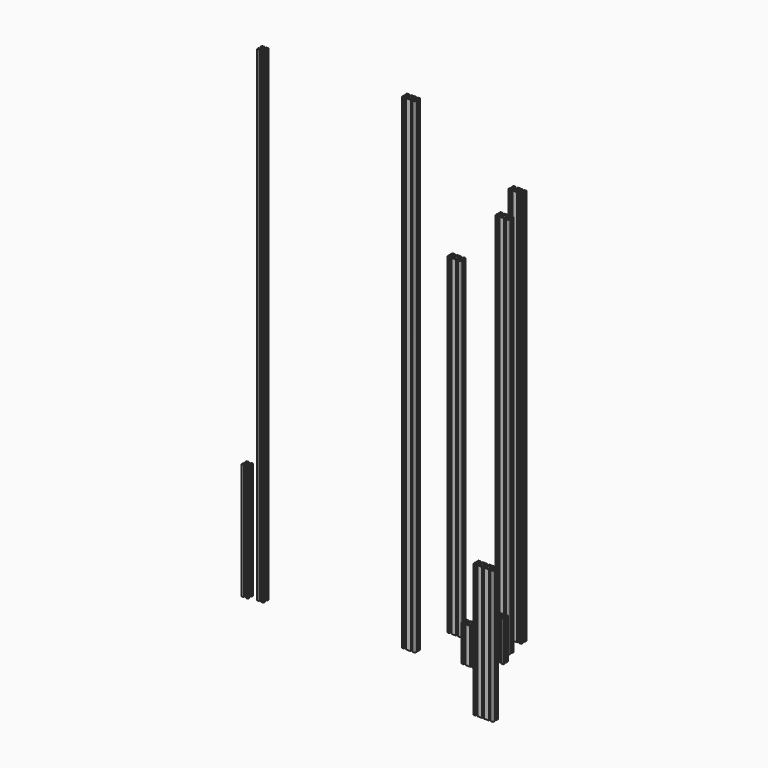
from build123d import *

# Parameters (mm, degrees)
F1_DEPTH  = 1192
F3_DEPTH  = 1152
F5_DEPTH  = 120
F7_DEPTH  = 1460
F9_DEPTH  = 108
F11_DEPTH = 400
F13_DEPTH = 996
F15_DEPTH = 350
F17_DEPTH = 1460


# Not quite as in the source:
# - ends of sketch curves that miss each other by under 0.0002 mm in the source are joined


with BuildPart() as f1:
    # F0 (on Top) → F1 (new body)
    with BuildSketch(Plane.XY):
        with BuildLine():
            ThreePointArc((1.538026356, 54.3189846685), (1.1788167823, 54.1701951914), (1.0300273052, 53.8109856177))
            Line((1.0300273052, 53.8109856177), (1.0300243052, 53.3269865693))
            ThreePointArc((1.0300243052, 53.3269865693), (1.1788167823, 52.9677769957), (1.538026356, 52.8189875185))
            Line((1.538026356, 52.8189875185), (6.9000258922, 52.8189875185))
            ThreePointArc((6.9000258922, 52.8189875185), (7.96068617, 53.2583273907), (8.4000260422, 54.3189876685))
            Line((8.4000260422, 54.3189876685), (8.4000260422, 59.6809872047))
            ThreePointArc((8.4000260422, 59.6809872047), (8.251236565, 60.0401967784), (7.8920269914, 60.1889862555))
            Line((7.8920269914, 60.1889862555), (7.408024943, 60.1889862555))
            ThreePointArc((7.408024943, 60.1889862555), (7.0488153693, 60.0401967784), (6.9000258922, 59.6809872047))
            Line((6.9000258922, 59.6809872047), (6.9000258922, 57.3319869698))
            ThreePointArc((6.9000258922, 57.3319869698), (6.751236415, 56.9727773962), (6.3920268414, 56.823987919))
            Line((6.3920268414, 56.823987919), (5.6661077688, 56.823987919))
            ThreePointArc((5.6661077688, 56.823987919), (5.4717049484, 56.8626570443), (5.3068981951, 56.9727773962))
            Line((5.3068981951, 56.9727773962), (2.2038164225, 60.0758562442))
            ThreePointArc((2.2038164225, 60.0758562442), (2.0936949388, 60.2406634798), (2.0550254077, 60.4350672802))
            Line((2.0550254077, 60.4350672802), (2.0550254077, 65.2029077569))
            ThreePointArc((2.0550254077, 65.2029077569), (2.0936949388, 65.3973115573), (2.2038163848, 65.5621188306))
            Line((2.2038163848, 65.5621188306), (5.3068967329, 68.6651991032))
            ThreePointArc((5.3068967329, 68.6651991032), (5.4717049484, 68.7753179928), (5.6661077688, 68.813987118))
            Line((5.6661077688, 68.813987118), (6.3920268414, 68.813987118))
            ThreePointArc((6.3920268414, 68.813987118), (6.751236415, 68.6651976409), (6.9000258922, 68.3059880672))
            Line((6.9000258922, 68.3059880672), (6.9000258922, 65.9569878323))
            ThreePointArc((6.9000258922, 65.9569878323), (7.0488153693, 65.5977782587), (7.408024943, 65.4489887815))
            Line((7.408024943, 65.4489887815), (7.8920269914, 65.4489887815))
            ThreePointArc((7.8920269914, 65.4489887815), (8.251236565, 65.5977782587), (8.4000260422, 65.9569878323))
            Line((8.4000260422, 65.9569878323), (8.4000260422, 71.3189873685))
            ThreePointArc((8.4000260422, 71.3189873685), (7.96068617, 72.3796476464), (6.9000258922, 72.8189875185))
            Line((6.9000258922, 72.8189875185), (1.538026356, 72.8189875185))
            ThreePointArc((1.538026356, 72.8189875185), (1.1788167823, 72.6701980414), (1.0300273052, 72.3109884677))
            Line((1.0300273052, 72.3109884677), (1.0300243052, 71.8269894193))
            ThreePointArc((1.0300243052, 71.8269894193), (1.1788167823, 71.4677798457), (1.538026356, 71.3189903685))
            Line((1.538026356, 71.3189903685), (3.8870265909, 71.3189873685))
            ThreePointArc((3.8870265909, 71.3189873685), (4.2462361645, 71.1701978914), (4.3950256417, 70.8109883177))
            Line((4.3950256417, 70.8109883177), (4.3950256417, 70.0850692452))
            ThreePointArc((4.3950256417, 70.0850692452), (4.3563561105, 69.8906654448), (4.2462346645, 69.7258581715))
            Line((4.2462346645, 69.7258581715), (1.1431543165, 66.6227778989))
            ThreePointArc((1.1431543165, 66.6227778989), (0.978346101, 66.5126590093), (0.7839432806, 66.473989884))
            Line((0.7839432806, 66.473989884), (-3.9838941962, 66.473986884))
            ThreePointArc((-3.9838941962, 66.473986884), (-4.1782970166, 66.5126590093), (-4.3431037699, 66.6227793612))
            Line((-4.3431037699, 66.6227793612), (-7.4461855425, 69.7258582092))
            ThreePointArc((-7.4461855425, 69.7258582092), (-7.5563044321, 69.8906664248), (-7.5949735573, 70.0850692452))
            Line((-7.5949735573, 70.0850692452), (-7.5949765573, 70.8109883177))
            ThreePointArc((-7.5949765573, 70.8109883177), (-7.4461840802, 71.1701978914), (-7.0869745065, 71.3189873685))
            Line((-7.0869745065, 71.3189873685), (-4.7379742716, 71.3189873685))
            ThreePointArc((-4.7379742716, 71.3189873685), (-4.378764698, 71.4677798457), (-4.2299752208, 71.8269894193))
            Line((-4.2299752208, 71.8269894193), (-4.2299752208, 72.3109884677))
            ThreePointArc((-4.2299752208, 72.3109884677), (-4.378764698, 72.6701980414), (-4.7379742716, 72.8189875185))
            Line((-4.7379742716, 72.8189875185), (-18.461976644, 72.8189875185))
            ThreePointArc((-18.461976644, 72.8189875185), (-18.8211862177, 72.6701980414), (-18.9699756948, 72.3109884677))
            Line((-18.9699756948, 72.3109884677), (-18.9699756948, 71.8269894193))
            ThreePointArc((-18.9699756948, 71.8269894193), (-18.8211862177, 71.4677798457), (-18.461976644, 71.3189903685))
            Line((-18.461976644, 71.3189903685), (-16.1129764091, 71.3189873685))
            ThreePointArc((-16.1129764091, 71.3189873685), (-15.7537668355, 71.1701978914), (-15.6049773583, 70.8109883177))
            Line((-15.6049773583, 70.8109883177), (-15.6049773583, 70.0850692452))
            ThreePointArc((-15.6049773583, 70.0850692452), (-15.6436464836, 69.8906664248), (-15.7537668355, 69.7258596715))
            Line((-15.7537668355, 69.7258596715), (-18.8568456835, 66.6227778989))
            ThreePointArc((-18.8568456835, 66.6227778989), (-19.021653899, 66.5126590093), (-19.2160567194, 66.473989884))
            Line((-19.2160567194, 66.473989884), (-23.9838971962, 66.473986884))
            ThreePointArc((-23.9838971962, 66.473986884), (-24.1783000166, 66.5126590093), (-24.3431067699, 66.6227793612))
            Line((-24.3431067699, 66.6227793612), (-27.4461885425, 69.7258582092))
            ThreePointArc((-27.4461885425, 69.7258582092), (-27.5563074321, 69.8906664248), (-27.5949765573, 70.0850692452))
            Line((-27.5949765573, 70.0850692452), (-27.5949765573, 70.8109883177))
            ThreePointArc((-27.5949765573, 70.8109883177), (-27.4461870802, 71.1701978914), (-27.0869775065, 71.3189873685))
            Line((-27.0869775065, 71.3189873685), (-24.7379772716, 71.3189873685))
            ThreePointArc((-24.7379772716, 71.3189873685), (-24.378767698, 71.4677798457), (-24.2299782208, 71.8269894193))
            Line((-24.2299782208, 71.8269894193), (-24.2299782208, 72.3109884677))
            ThreePointArc((-24.2299782208, 72.3109884677), (-24.378767698, 72.6701980414), (-24.7379772716, 72.8189875185))
            Line((-24.7379772716, 72.8189875185), (-30.0999768078, 72.8189875185))
            ThreePointArc((-30.0999768078, 72.8189875185), (-31.1606370857, 72.3796476464), (-31.5999769578, 71.3189873685))
            Line((-31.5999769578, 71.3189873685), (-31.5999769578, 65.9569878323))
            ThreePointArc((-31.5999769578, 65.9569878323), (-31.4511874807, 65.5977782587), (-31.091977907, 65.4489887815))
            Line((-31.091977907, 65.4489887815), (-30.6079788586, 65.4489887815))
            ThreePointArc((-30.6079788586, 65.4489887815), (-30.248769285, 65.5977782587), (-30.0999798078, 65.9569878323))
            Line((-30.0999798078, 65.9569878323), (-30.0999768078, 68.3059880672))
            ThreePointArc((-30.0999768078, 68.3059880672), (-29.9511873307, 68.6651976409), (-29.591977757, 68.813987118))
            Line((-29.591977757, 68.813987118), (-28.8660586844, 68.813987118))
            ThreePointArc((-28.8660586844, 68.813987118), (-28.671655864, 68.7753179928), (-28.5068491108, 68.6651976409))
            Line((-28.5068491108, 68.6651976409), (-25.4037673382, 65.5621187929))
            ThreePointArc((-25.4037673382, 65.5621187929), (-25.2936484486, 65.3973105773), (-25.2549793233, 65.2029077569))
            Line((-25.2549793233, 65.2029077569), (-25.2549763233, 60.4350672802))
            ThreePointArc((-25.2549763233, 60.4350672802), (-25.2936484486, 60.2406644598), (-25.4037688005, 60.0758577065))
            Line((-25.4037688005, 60.0758577065), (-28.5068476485, 56.9727759339))
            ThreePointArc((-28.5068476485, 56.9727759339), (-28.671655864, 56.8626570443), (-28.8660586844, 56.823987919))
            Line((-28.8660586844, 56.823987919), (-29.591977757, 56.823987919))
            ThreePointArc((-29.591977757, 56.823987919), (-29.9511873307, 56.9727773962), (-30.0999768078, 57.3319869698))
            Line((-30.0999768078, 57.3319869698), (-30.0999768078, 59.6809872047))
            ThreePointArc((-30.0999768078, 59.6809872047), (-30.248769285, 60.0401967784), (-30.6079788586, 60.1889862555))
            Line((-30.6079788586, 60.1889862555), (-31.091977907, 60.1889862555))
            ThreePointArc((-31.091977907, 60.1889862555), (-31.4511874807, 60.0401967784), (-31.5999769578, 59.6809872047))
            Line((-31.5999769578, 59.6809872047), (-31.5999769578, 54.3189876685))
            ThreePointArc((-31.5999769578, 54.3189876685), (-31.1606370857, 53.2583273907), (-30.0999768078, 52.8189875185))
            Line((-30.0999768078, 52.8189875185), (-24.7379772716, 52.8189875185))
            ThreePointArc((-24.7379772716, 52.8189875185), (-24.378767698, 52.9677769957), (-24.2299782208, 53.3269865693))
            Line((-24.2299782208, 53.3269865693), (-24.2299782208, 53.8109856177))
            ThreePointArc((-24.2299782208, 53.8109856177), (-24.378767698, 54.1701951914), (-24.7379772716, 54.3189846685))
            Line((-24.7379772716, 54.3189846685), (-27.0869775065, 54.3189876685))
            ThreePointArc((-27.0869775065, 54.3189876685), (-27.4461870802, 54.4677771457), (-27.5949765573, 54.8269867193))
            Line((-27.5949765573, 54.8269867193), (-27.5949765573, 55.5529057919))
            ThreePointArc((-27.5949765573, 55.5529057919), (-27.5563074321, 55.7473086123), (-27.4461870802, 55.9121153656))
            Line((-27.4461870802, 55.9121153656), (-24.3431082321, 59.0151971382))
            ThreePointArc((-24.3431082321, 59.0151971382), (-24.1783000166, 59.1253160278), (-23.9838971962, 59.163985153))
            Line((-23.9838971962, 59.163985153), (-19.2160567194, 59.163988153))
            ThreePointArc((-19.2160567194, 59.163988153), (-19.021653899, 59.1253160278), (-18.8568471458, 59.0151956759))
            Line((-18.8568471458, 59.0151956759), (-15.7537653732, 55.9121168279))
            ThreePointArc((-15.7537653732, 55.9121168279), (-15.6436464836, 55.7473086123), (-15.6049773583, 55.5529057919))
            Line((-15.6049773583, 55.5529057919), (-15.6049773583, 54.8269867193))
            ThreePointArc((-15.6049773583, 54.8269867193), (-15.7537668355, 54.4677771457), (-16.1129764091, 54.3189876685))
            Line((-16.1129764091, 54.3189876685), (-18.461976644, 54.3189876685))
            ThreePointArc((-18.461976644, 54.3189876685), (-18.8211862177, 54.1701951914), (-18.9699756948, 53.8109856177))
            Line((-18.9699756948, 53.8109856177), (-18.9699756948, 53.3269865693))
            ThreePointArc((-18.9699756948, 53.3269865693), (-18.8211862177, 52.9677769957), (-18.461976644, 52.8189875185))
            Line((-18.461976644, 52.8189875185), (-4.7379742716, 52.8189875185))
            ThreePointArc((-4.7379742716, 52.8189875185), (-4.378764698, 52.9677769957), (-4.2299752208, 53.3269865693))
            Line((-4.2299752208, 53.3269865693), (-4.2299752208, 53.8109856177))
            ThreePointArc((-4.2299752208, 53.8109856177), (-4.378764698, 54.1701951914), (-4.7379742716, 54.3189846685))
            Line((-4.7379742716, 54.3189846685), (-7.0869745065, 54.3189876685))
            ThreePointArc((-7.0869745065, 54.3189876685), (-7.4461840802, 54.4677771457), (-7.5949735573, 54.8269867193))
            Line((-7.5949735573, 54.8269867193), (-7.5949765573, 55.5529057919))
            ThreePointArc((-7.5949765573, 55.5529057919), (-7.5563044321, 55.7473086123), (-7.4461840802, 55.9121153656))
            Line((-7.4461840802, 55.9121153656), (-4.3431052321, 59.0151971382))
            ThreePointArc((-4.3431052321, 59.0151971382), (-4.1782970166, 59.1253160278), (-3.9838941962, 59.163985153))
            Line((-3.9838941962, 59.163985153), (0.7839432806, 59.163988153))
            ThreePointArc((0.7839432806, 59.163988153), (0.978346101, 59.1253160278), (1.1431528542, 59.0151956759))
            Line((1.1431528542, 59.0151956759), (4.2462346268, 55.9121168279))
            ThreePointArc((4.2462346268, 55.9121168279), (4.3563561105, 55.7473095923), (4.3950256417, 55.5529057919))
            Line((4.3950256417, 55.5529057919), (4.3950256417, 54.8269867193))
            ThreePointArc((4.3950256417, 54.8269867193), (4.2462361645, 54.4677771457), (3.8870265909, 54.3189876685))
            Line((3.8870265909, 54.3189876685), (1.538026356, 54.3189846685))
        make_face()
        with BuildLine():
            ThreePointArc((-20.7959977744, 64.7541219525), (-20.2435081236, 65.3249247328), (-19.4750769157, 65.1234945787))
            Line((-19.4750769157, 65.1234945787), (-19.2954697274, 64.943887731))
            ThreePointArc((-19.2954697274, 64.943887731), (-19.0940397436, 64.1754563528), (-19.6648425239, 63.622966702))
            ThreePointArc((-19.6648425239, 63.622966702), (-19.5044767483, 62.8189875185), (-19.6648427838, 62.0150118617))
            ThreePointArc((-19.6648427838, 62.0150118617), (-19.0940397436, 61.4625186843), (-19.2954698977, 60.6940874764))
            Line((-19.2954698977, 60.6940874764), (-19.4750767453, 60.5144802881))
            ThreePointArc((-19.4750767453, 60.5144802881), (-20.2435081236, 60.3130503043), (-20.7959977744, 60.8838530846))
            ThreePointArc((-20.7959977744, 60.8838530846), (-21.5999769578, 60.723487309), (-22.4039526147, 60.8838533445))
            ThreePointArc((-22.4039526147, 60.8838533445), (-22.9564457921, 60.3130503043), (-23.724877, 60.5144804584))
            Line((-23.724877, 60.5144804584), (-23.9044841883, 60.6940873061))
            ThreePointArc((-23.9044841883, 60.6940873061), (-24.1059141721, 61.4625186843), (-23.5351113918, 62.0150083351))
            ThreePointArc((-23.5351113918, 62.0150083351), (-23.6954771674, 62.8189875185), (-23.5351111318, 63.6229631754))
            ThreePointArc((-23.5351111318, 63.6229631754), (-24.1059141721, 64.1754563528), (-23.904484018, 64.9438875607))
            Line((-23.904484018, 64.9438875607), (-23.7248771703, 65.123494749))
            ThreePointArc((-23.7248771703, 65.123494749), (-22.9564457921, 65.3249247328), (-22.4039561413, 64.7541219525))
            ThreePointArc((-22.4039561413, 64.7541219525), (-21.5999769578, 64.9144877281), (-20.7959977744, 64.7541219525))
        make_face(mode=Mode.SUBTRACT)
        with BuildLine():
            ThreePointArc((-5.4037658005, 65.5621173306), (-5.2936454486, 65.3973105773), (-5.2549763233, 65.2029077569))
            Line((-5.2549763233, 65.2029077569), (-5.2549763233, 60.4350672802))
            ThreePointArc((-5.2549763233, 60.4350672802), (-5.2936454486, 60.2406644598), (-5.4037658005, 60.0758577065))
            Line((-5.4037658005, 60.0758577065), (-8.9461856925, 56.53343789))
            ThreePointArc((-8.9461856925, 56.53343789), (-9.0563045821, 56.3686296745), (-9.0949737073, 56.1742268541))
            Line((-9.0949737073, 56.1742268541), (-9.0949767073, 54.8269867193))
            ThreePointArc((-9.0949767073, 54.8269867193), (-9.2437661845, 54.4677771457), (-9.6029757581, 54.3189876685))
            Line((-9.6029757581, 54.3189876685), (-13.5969751575, 54.3189876685))
            ThreePointArc((-13.5969751575, 54.3189876685), (-13.9561847312, 54.4677771457), (-14.1049742083, 54.8269867193))
            Line((-14.1049742083, 54.8269867193), (-14.1049772083, 56.1742268541))
            ThreePointArc((-14.1049772083, 56.1742268541), (-14.1436463336, 56.3686296745), (-14.2537666855, 56.5334364277))
            Line((-14.2537666855, 56.5334364277), (-17.7961865775, 60.0758562442))
            ThreePointArc((-17.7961865775, 60.0758562442), (-17.9063054671, 60.2406644598), (-17.9449745923, 60.4350672802))
            Line((-17.9449745923, 60.4350672802), (-17.9449775923, 65.2029077569))
            ThreePointArc((-17.9449775923, 65.2029077569), (-17.9063054671, 65.3973105773), (-17.7961851152, 65.5621173306))
            Line((-17.7961851152, 65.5621173306), (-14.2537652232, 69.1045371471))
            ThreePointArc((-14.2537652232, 69.1045371471), (-14.1436463336, 69.2693453626), (-14.1049772083, 69.463748183))
            Line((-14.1049772083, 69.463748183), (-14.1049772083, 70.8109883177))
            ThreePointArc((-14.1049772083, 70.8109883177), (-13.9561847312, 71.1701978914), (-13.5969751575, 71.3189873685))
            Line((-13.5969751575, 71.3189873685), (-9.6029757581, 71.3189873685))
            ThreePointArc((-9.6029757581, 71.3189873685), (-9.2437661845, 71.1701978914), (-9.0949767073, 70.8109883177))
            Line((-9.0949767073, 70.8109883177), (-9.0949767073, 69.463748183))
            ThreePointArc((-9.0949767073, 69.463748183), (-9.0563045821, 69.2693453626), (-8.9461842302, 69.1045386094))
            Line((-8.9461842302, 69.1045386094), (-5.4037658005, 65.5621173306))
        make_face(mode=Mode.SUBTRACT)
        with BuildLine():
            ThreePointArc((-2.4039521731, 64.7541206296), (-1.599975343, 64.9144877281), (-0.795998301, 64.7541216926))
            ThreePointArc((-0.795998301, 64.7541216926), (-0.2435067586, 65.3249251145), (0.5249245843, 65.1234930787))
            Line((0.5249245843, 65.1234930787), (0.7045302726, 64.943887731))
            ThreePointArc((0.7045302726, 64.943887731), (0.9059631497, 64.1754559711), (0.3351576457, 63.6229660091))
            ThreePointArc((0.3351576457, 63.6229660091), (0.4955262517, 62.8189875185), (0.3351597746, 62.0150107988))
            ThreePointArc((0.3351597746, 62.0150107988), (0.9059631497, 61.462519066), (0.7045316023, 60.6940859764))
            Line((0.7045316023, 60.6940859764), (0.5249262547, 60.5144802881))
            ThreePointArc((0.5249262547, 60.5144802881), (-0.2435067586, 60.3130499226), (-0.7959976048, 60.8838523918))
            ThreePointArc((-0.7959976048, 60.8838523918), (-1.599975343, 60.723487309), (-2.4039521731, 60.8838544075))
            ThreePointArc((-2.4039521731, 60.8838544075), (-2.956444157, 60.3130499226), (-3.7248755, 60.5144819584))
            Line((-3.7248755, 60.5144819584), (-3.9044811883, 60.6940873061))
            ThreePointArc((-3.9044811883, 60.6940873061), (-4.1059111721, 61.4625186843), (-3.5351083918, 62.0150083351))
            ThreePointArc((-3.5351083918, 62.0150083351), (-3.6954741674, 62.8189875185), (-3.5351081318, 63.6229631754))
            ThreePointArc((-3.5351081318, 63.6229631754), (-4.1059111721, 64.1754563528), (-3.904481018, 64.9438875607))
            Line((-3.904481018, 64.9438875607), (-3.7248771703, 65.123494749))
            ThreePointArc((-3.7248771703, 65.123494749), (-2.956444157, 65.3249251145), (-2.4039521731, 64.7541206296))
        make_face(mode=Mode.SUBTRACT)
    extrude(amount=F1_DEPTH)


with BuildPart() as f3:
    # F2 (on Top) → F3 (new body)
    with BuildSketch(Plane.XY):
        with BuildLine():
            ThreePointArc((13.1380145138, -8.50000285), (12.7788049401, -8.6487923271), (12.630015463, -9.0080019008))
            Line((12.630015463, -9.0080019008), (12.630012463, -9.4920009492))
            ThreePointArc((12.630012463, -9.4920009492), (12.7788049401, -9.8512105229), (13.1380145138, -10))
            Line((13.1380145138, -10), (18.50001405, -10))
            ThreePointArc((18.50001405, -10), (19.5606743278, -9.5606601278), (20.0000142, -8.49999985))
            Line((20.0000142, -8.49999985), (20.0000142, -3.1380003138))
            ThreePointArc((20.0000142, -3.1380003138), (19.8512247229, -2.7787907401), (19.4920151492, -2.630001263))
            Line((19.4920151492, -2.630001263), (19.0080131008, -2.630001263))
            ThreePointArc((19.0080131008, -2.630001263), (18.6488035271, -2.7787907401), (18.50001405, -3.1380003138))
            Line((18.50001405, -3.1380003138), (18.50001405, -5.4870005487))
            ThreePointArc((18.50001405, -5.4870005487), (18.3512245729, -5.8462101224), (17.9920149992, -5.9949995995))
            Line((17.9920149992, -5.9949995995), (17.2660959266, -5.9949995995))
            ThreePointArc((17.2660959266, -5.9949995995), (17.0716931062, -5.9563304743), (16.906886353, -5.8462101224))
            Line((16.906886353, -5.8462101224), (13.8038045804, -2.7431312743))
            ThreePointArc((13.8038045804, -2.7431312743), (13.6936830966, -2.5783240387), (13.6550135655, -2.3839202384))
            Line((13.6550135655, -2.3839202384), (13.6550135655, 2.3839202384))
            ThreePointArc((13.6550135655, 2.3839202384), (13.6936830966, 2.5783240387), (13.8038045426, 2.743131312))
            Line((13.8038045426, 2.743131312), (16.9068848907, 5.8462115846))
            ThreePointArc((16.9068848907, 5.8462115846), (17.0716931062, 5.9563304743), (17.2660959266, 5.9949995995))
            Line((17.2660959266, 5.9949995995), (17.9920149992, 5.9949995995))
            ThreePointArc((17.9920149992, 5.9949995995), (18.3512245729, 5.8462101224), (18.50001405, 5.4870005487))
            Line((18.50001405, 5.4870005487), (18.50001405, 3.1380003138))
            ThreePointArc((18.50001405, 3.1380003138), (18.6488035271, 2.7787907401), (19.0080131008, 2.630001263))
            Line((19.0080131008, 2.630001263), (19.4920151492, 2.630001263))
            ThreePointArc((19.4920151492, 2.630001263), (19.8512247229, 2.7787907401), (20.0000142, 3.1380003138))
            Line((20.0000142, 3.1380003138), (20.0000142, 8.49999985))
            ThreePointArc((20.0000142, 8.49999985), (19.5606743278, 9.5606601278), (18.50001405, 10))
            Line((18.50001405, 10), (13.1380145138, 10))
            ThreePointArc((13.1380145138, 10), (12.7788049401, 9.8512105229), (12.630015463, 9.4920009492))
            Line((12.630015463, 9.4920009492), (12.630012463, 9.0080019008))
            ThreePointArc((12.630012463, 9.0080019008), (12.7788049401, 8.6487923271), (13.1380145138, 8.50000285))
            Line((13.1380145138, 8.50000285), (15.4870147487, 8.49999985))
            ThreePointArc((15.4870147487, 8.49999985), (15.8462243224, 8.3512103729), (15.9950137995, 7.9920007992))
            Line((15.9950137995, 7.9920007992), (15.9950137995, 7.2660817266))
            ThreePointArc((15.9950137995, 7.2660817266), (15.9563442684, 7.0716779263), (15.8462228224, 6.906870653))
            Line((15.8462228224, 6.906870653), (12.7431424743, 3.8037903804))
            ThreePointArc((12.7431424743, 3.8037903804), (12.5783342588, 3.6936714907), (12.3839314384, 3.6550023655))
            Line((12.3839314384, 3.6550023655), (7.6160939616, 3.6549993655))
            ThreePointArc((7.6160939616, 3.6549993655), (7.4216911412, 3.6936714907), (7.256884388, 3.8037918426))
            Line((7.256884388, 3.8037918426), (4.1538026154, 6.9068706907))
            ThreePointArc((4.1538026154, 6.9068706907), (4.0436837257, 7.0716789062), (4.0050146005, 7.2660817266))
            Line((4.0050146005, 7.2660817266), (4.0050116005, 7.9920007992))
            ThreePointArc((4.0050116005, 7.9920007992), (4.1538040776, 8.3512103729), (4.5130136513, 8.49999985))
            Line((4.5130136513, 8.49999985), (6.8620138862, 8.49999985))
            ThreePointArc((6.8620138862, 8.49999985), (7.2212234599, 8.6487923271), (7.370012937, 9.0080019008))
            Line((7.370012937, 9.0080019008), (7.370012937, 9.4920009492))
            ThreePointArc((7.370012937, 9.4920009492), (7.2212234599, 9.8512105229), (6.8620138862, 10))
            Line((6.8620138862, 10), (-6.8619884862, 10))
            ThreePointArc((-6.8619884862, 10), (-7.2211980599, 9.8512105229), (-7.369987537, 9.4920009492))
            Line((-7.369987537, 9.4920009492), (-7.369987537, 9.0080019008))
            ThreePointArc((-7.369987537, 9.0080019008), (-7.2211980599, 8.6487923271), (-6.8619884862, 8.50000285))
            Line((-6.8619884862, 8.50000285), (-4.5129882513, 8.49999985))
            ThreePointArc((-4.5129882513, 8.49999985), (-4.1537786776, 8.3512103729), (-4.0049892005, 7.9920007992))
            Line((-4.0049892005, 7.9920007992), (-4.0049892005, 7.2660817266))
            ThreePointArc((-4.0049892005, 7.2660817266), (-4.0436583257, 7.0716789062), (-4.1537786776, 6.906872153))
            Line((-4.1537786776, 6.906872153), (-7.2568575257, 3.8037903804))
            ThreePointArc((-7.2568575257, 3.8037903804), (-7.4216657412, 3.6936714907), (-7.6160685616, 3.6550023655))
            Line((-7.6160685616, 3.6550023655), (-12.3839090384, 3.6549993655))
            ThreePointArc((-12.3839090384, 3.6549993655), (-12.5783118588, 3.6936714907), (-12.743118612, 3.8037918426))
            Line((-12.743118612, 3.8037918426), (-15.8462003846, 6.9068706907))
            ThreePointArc((-15.8462003846, 6.9068706907), (-15.9563192743, 7.0716789062), (-15.9949883995, 7.2660817266))
            Line((-15.9949883995, 7.2660817266), (-15.9949883995, 7.9920007992))
            ThreePointArc((-15.9949883995, 7.9920007992), (-15.8461989224, 8.3512103729), (-15.4869893487, 8.49999985))
            Line((-15.4869893487, 8.49999985), (-13.1379891138, 8.49999985))
            ThreePointArc((-13.1379891138, 8.49999985), (-12.7787795401, 8.6487923271), (-12.629990063, 9.0080019008))
            Line((-12.629990063, 9.0080019008), (-12.629990063, 9.4920009492))
            ThreePointArc((-12.629990063, 9.4920009492), (-12.7787795401, 9.8512105229), (-13.1379891138, 10))
            Line((-13.1379891138, 10), (-18.49998865, 10))
            ThreePointArc((-18.49998865, 10), (-19.5606489278, 9.5606601278), (-19.9999888, 8.49999985))
            Line((-19.9999888, 8.49999985), (-19.9999888, 3.1380003138))
            ThreePointArc((-19.9999888, 3.1380003138), (-19.8511993229, 2.7787907401), (-19.4919897492, 2.630001263))
            Line((-19.4919897492, 2.630001263), (-19.0079907008, 2.630001263))
            ThreePointArc((-19.0079907008, 2.630001263), (-18.6487811271, 2.7787907401), (-18.49999165, 3.1380003138))
            Line((-18.49999165, 3.1380003138), (-18.49998865, 5.4870005487))
            ThreePointArc((-18.49998865, 5.4870005487), (-18.3511991729, 5.8462101224), (-17.9919895992, 5.9949995995))
            Line((-17.9919895992, 5.9949995995), (-17.2660705266, 5.9949995995))
            ThreePointArc((-17.2660705266, 5.9949995995), (-17.0716677062, 5.9563304743), (-16.906860953, 5.8462101224))
            Line((-16.906860953, 5.8462101224), (-13.8037791804, 2.7431312743))
            ThreePointArc((-13.8037791804, 2.7431312743), (-13.6936602907, 2.5783230588), (-13.6549911655, 2.3839202384))
            Line((-13.6549911655, 2.3839202384), (-13.6549881655, -2.3839202384))
            ThreePointArc((-13.6549881655, -2.3839202384), (-13.6936602907, -2.5783230588), (-13.8037806426, -2.743129812))
            Line((-13.8037806426, -2.743129812), (-16.9068594907, -5.8462115846))
            ThreePointArc((-16.9068594907, -5.8462115846), (-17.0716677062, -5.9563304743), (-17.2660705266, -5.9949995995))
            Line((-17.2660705266, -5.9949995995), (-17.9919895992, -5.9949995995))
            ThreePointArc((-17.9919895992, -5.9949995995), (-18.3511991729, -5.8462101224), (-18.49998865, -5.4870005487))
            Line((-18.49998865, -5.4870005487), (-18.49998865, -3.1380003138))
            ThreePointArc((-18.49998865, -3.1380003138), (-18.6487811271, -2.7787907401), (-19.0079907008, -2.630001263))
            Line((-19.0079907008, -2.630001263), (-19.4919897492, -2.630001263))
            ThreePointArc((-19.4919897492, -2.630001263), (-19.8511993229, -2.7787907401), (-19.9999888, -3.1380003138))
            Line((-19.9999888, -3.1380003138), (-19.9999888, -8.49999985))
            ThreePointArc((-19.9999888, -8.49999985), (-19.5606489278, -9.5606601278), (-18.49998865, -10))
            Line((-18.49998865, -10), (-13.1379891138, -10))
            ThreePointArc((-13.1379891138, -10), (-12.7787795401, -9.8512105229), (-12.629990063, -9.4920009492))
            Line((-12.629990063, -9.4920009492), (-12.629990063, -9.0080019008))
            ThreePointArc((-12.629990063, -9.0080019008), (-12.7787795401, -8.6487923271), (-13.1379891138, -8.50000285))
            Line((-13.1379891138, -8.50000285), (-15.4869893487, -8.49999985))
            ThreePointArc((-15.4869893487, -8.49999985), (-15.8461989224, -8.3512103729), (-15.9949883995, -7.9920007992))
            Line((-15.9949883995, -7.9920007992), (-15.9949883995, -7.2660817266))
            ThreePointArc((-15.9949883995, -7.2660817266), (-15.9563192743, -7.0716789062), (-15.8461989224, -6.906872153))
            Line((-15.8461989224, -6.906872153), (-12.7431200743, -3.8037903804))
            ThreePointArc((-12.7431200743, -3.8037903804), (-12.5783118588, -3.6936714907), (-12.3839090384, -3.6550023655))
            Line((-12.3839090384, -3.6550023655), (-7.6160685616, -3.6549993655))
            ThreePointArc((-7.6160685616, -3.6549993655), (-7.4216657412, -3.6936714907), (-7.256858988, -3.8037918426))
            Line((-7.256858988, -3.8037918426), (-4.1537772154, -6.9068706907))
            ThreePointArc((-4.1537772154, -6.9068706907), (-4.0436583257, -7.0716789062), (-4.0049892005, -7.2660817266))
            Line((-4.0049892005, -7.2660817266), (-4.0049892005, -7.9920007992))
            ThreePointArc((-4.0049892005, -7.9920007992), (-4.1537786776, -8.3512103729), (-4.5129882513, -8.49999985))
            Line((-4.5129882513, -8.49999985), (-6.8619884862, -8.49999985))
            ThreePointArc((-6.8619884862, -8.49999985), (-7.2211980599, -8.6487923271), (-7.369987537, -9.0080019008))
            Line((-7.369987537, -9.0080019008), (-7.369987537, -9.4920009492))
            ThreePointArc((-7.369987537, -9.4920009492), (-7.2211980599, -9.8512105229), (-6.8619884862, -10))
            Line((-6.8619884862, -10), (6.8620138862, -10))
            ThreePointArc((6.8620138862, -10), (7.2212234599, -9.8512105229), (7.370012937, -9.4920009492))
            Line((7.370012937, -9.4920009492), (7.370012937, -9.0080019008))
            ThreePointArc((7.370012937, -9.0080019008), (7.2212234599, -8.6487923271), (6.8620138862, -8.50000285))
            Line((6.8620138862, -8.50000285), (4.5130136513, -8.49999985))
            ThreePointArc((4.5130136513, -8.49999985), (4.1538040776, -8.3512103729), (4.0050146005, -7.9920007992))
            Line((4.0050146005, -7.9920007992), (4.0050116005, -7.2660817266))
            ThreePointArc((4.0050116005, -7.2660817266), (4.0436837257, -7.0716789062), (4.1538040776, -6.906872153))
            Line((4.1538040776, -6.906872153), (7.2568829257, -3.8037903804))
            ThreePointArc((7.2568829257, -3.8037903804), (7.4216911412, -3.6936714907), (7.6160939616, -3.6550023655))
            Line((7.6160939616, -3.6550023655), (12.3839314384, -3.6549993655))
            ThreePointArc((12.3839314384, -3.6549993655), (12.5783342588, -3.6936714907), (12.743141012, -3.8037918426))
            Line((12.743141012, -3.8037918426), (15.8462227846, -6.9068706907))
            ThreePointArc((15.8462227846, -6.9068706907), (15.9563442684, -7.0716779263), (15.9950137995, -7.2660817266))
            Line((15.9950137995, -7.2660817266), (15.9950137995, -7.9920007992))
            ThreePointArc((15.9950137995, -7.9920007992), (15.8462243224, -8.3512103729), (15.4870147487, -8.49999985))
            Line((15.4870147487, -8.49999985), (13.1380145138, -8.50000285))
        make_face()
        with BuildLine():
            ThreePointArc((-9.1960096166, 1.9351344339), (-8.6435199657, 2.5059372142), (-7.8750887578, 2.3045070601))
            Line((-7.8750887578, 2.3045070601), (-7.6954815695, 2.1249002125))
            ThreePointArc((-7.6954815695, 2.1249002125), (-7.4940515858, 1.3564688343), (-8.0648543661, 0.8039791834))
            ThreePointArc((-8.0648543661, 0.8039791834), (-7.9044885905, 0), (-8.064854626, -0.8039756568))
            ThreePointArc((-8.064854626, -0.8039756568), (-7.4940515858, -1.3564688343), (-7.6954817399, -2.1249000422))
            Line((-7.6954817399, -2.1249000422), (-7.8750885875, -2.3045072305))
            ThreePointArc((-7.8750885875, -2.3045072305), (-8.6435199657, -2.5059372142), (-9.1960096166, -1.9351344339))
            ThreePointArc((-9.1960096166, -1.9351344339), (-9.9999888, -2.0955002096), (-10.8039644568, -1.935134174))
            ThreePointArc((-10.8039644568, -1.935134174), (-11.3564576343, -2.5059372142), (-12.1248888422, -2.3045070601))
            Line((-12.1248888422, -2.3045070601), (-12.3044960305, -2.1249002125))
            ThreePointArc((-12.3044960305, -2.1249002125), (-12.5059260142, -1.3564688343), (-11.9351232339, -0.8039791834))
            ThreePointArc((-11.9351232339, -0.8039791834), (-12.0954890096, 0), (-11.935122974, 0.8039756568))
            ThreePointArc((-11.935122974, 0.8039756568), (-12.5059260142, 1.3564688343), (-12.3044958601, 2.1249000422))
            Line((-12.3044958601, 2.1249000422), (-12.1248890125, 2.3045072305))
            ThreePointArc((-12.1248890125, 2.3045072305), (-11.3564576343, 2.5059372142), (-10.8039679834, 1.9351344339))
            ThreePointArc((-10.8039679834, 1.9351344339), (-9.9999888, 2.0955002096), (-9.1960096166, 1.9351344339))
        make_face(mode=Mode.SUBTRACT)
        with BuildLine():
            ThreePointArc((6.1962223574, 2.743129812), (6.3063427093, 2.5783230588), (6.3450118345, 2.3839202384))
            Line((6.3450118345, 2.3839202384), (6.3450118345, -2.3839202384))
            ThreePointArc((6.3450118345, -2.3839202384), (6.3063427093, -2.5783230588), (6.1962223574, -2.743129812))
            Line((6.1962223574, -2.743129812), (2.6538024654, -6.2855496286))
            ThreePointArc((2.6538024654, -6.2855496286), (2.5436835757, -6.4503578441), (2.5050144505, -6.6447606645))
            Line((2.5050144505, -6.6447606645), (2.5050114505, -7.9920007992))
            ThreePointArc((2.5050114505, -7.9920007992), (2.3562219734, -8.3512103729), (1.9970123997, -8.49999985))
            Line((1.9970123997, -8.49999985), (-1.9969869997, -8.49999985))
            ThreePointArc((-1.9969869997, -8.49999985), (-2.3561965734, -8.3512103729), (-2.5049860505, -7.9920007992))
            Line((-2.5049860505, -7.9920007992), (-2.5049890505, -6.6447606645))
            ThreePointArc((-2.5049890505, -6.6447606645), (-2.5436581757, -6.4503578441), (-2.6537785276, -6.2855510908))
            Line((-2.6537785276, -6.2855510908), (-6.1961984196, -2.7431312743))
            ThreePointArc((-6.1961984196, -2.7431312743), (-6.3063173093, -2.5783230588), (-6.3449864345, -2.3839202384))
            Line((-6.3449864345, -2.3839202384), (-6.3449894345, 2.3839202384))
            ThreePointArc((-6.3449894345, 2.3839202384), (-6.3063173093, 2.5783230588), (-6.1961969574, 2.743129812))
            Line((-6.1961969574, 2.743129812), (-2.6537770654, 6.2855496286))
            ThreePointArc((-2.6537770654, 6.2855496286), (-2.5436581757, 6.4503578441), (-2.5049890505, 6.6447606645))
            Line((-2.5049890505, 6.6447606645), (-2.5049890505, 7.9920007992))
            ThreePointArc((-2.5049890505, 7.9920007992), (-2.3561965734, 8.3512103729), (-1.9969869997, 8.49999985))
            Line((-1.9969869997, 8.49999985), (1.9970123997, 8.49999985))
            ThreePointArc((1.9970123997, 8.49999985), (2.3562219734, 8.3512103729), (2.5050114505, 7.9920007992))
            Line((2.5050114505, 7.9920007992), (2.5050114505, 6.6447606645))
            ThreePointArc((2.5050114505, 6.6447606645), (2.5436835757, 6.4503578441), (2.6538039276, 6.2855510908))
            Line((2.6538039276, 6.2855510908), (6.1962223574, 2.743129812))
        make_face(mode=Mode.SUBTRACT)
        with BuildLine():
            ThreePointArc((9.1960359848, 1.9351331111), (10.0000128148, 2.0955002095), (10.8039898568, 1.935134174))
            ThreePointArc((10.8039898568, 1.935134174), (11.3564813992, 2.5059375959), (12.1249127422, 2.3045055601))
            Line((12.1249127422, 2.3045055601), (12.3045184305, 2.1249002125))
            ThreePointArc((12.3045184305, 2.1249002125), (12.5059513075, 1.3564684526), (11.9351458035, 0.8039784906))
            ThreePointArc((11.9351458035, 0.8039784906), (12.0955144096, 0), (11.9351479324, -0.8039767198))
            ThreePointArc((11.9351479324, -0.8039767198), (12.5059513075, -1.3564684526), (12.3045197601, -2.1249015422))
            Line((12.3045197601, -2.1249015422), (12.1249144125, -2.3045072305))
            ThreePointArc((12.1249144125, -2.3045072305), (11.3564813992, -2.5059375959), (10.803990553, -1.9351351268))
            ThreePointArc((10.803990553, -1.9351351268), (10.0000128148, -2.0955002095), (9.1960359848, -1.9351331111))
            ThreePointArc((9.1960359848, -1.9351331111), (8.6435440008, -2.5059375959), (7.8751126578, -2.3045055601))
            Line((7.8751126578, -2.3045055601), (7.6955069695, -2.1249002125))
            ThreePointArc((7.6955069695, -2.1249002125), (7.4940769858, -1.3564688343), (8.0648797661, -0.8039791834))
            ThreePointArc((8.0648797661, -0.8039791834), (7.9045139905, 0), (8.064880026, 0.8039756568))
            ThreePointArc((8.064880026, 0.8039756568), (7.4940769858, 1.3564688343), (7.6955071399, 2.1249000422))
            Line((7.6955071399, 2.1249000422), (7.8751109875, 2.3045072305))
            ThreePointArc((7.8751109875, 2.3045072305), (8.6435440008, 2.5059375959), (9.1960359848, 1.9351331111))
        make_face(mode=Mode.SUBTRACT)
    extrude(amount=F3_DEPTH)


with BuildPart() as f5:
    # F4 (on Top) → F5 (new body)
    with BuildSketch(Plane.XY):
        with BuildLine():
            ThreePointArc((-6.8620003529, -53.6000005195), (-7.2212099265, -53.7487899966), (-7.3699994037, -54.1079995703))
            Line((-7.3699994037, -54.1079995703), (-7.3700024037, -54.5919986187))
            ThreePointArc((-7.3700024037, -54.5919986187), (-7.2212099265, -54.9512081923), (-6.8620003529, -55.0999976695))
            Line((-6.8620003529, -55.0999976695), (-1.5000008167, -55.0999976695))
            Line((-1.5000008167, -55.0999976695), (6.8619990195, -55.0999976695))
            ThreePointArc((6.8619990195, -55.0999976695), (7.2212085932, -54.9512081923), (7.3699980703, -54.5919986187))
            Line((7.3699980703, -54.5919986187), (7.3700010703, -54.1079995703))
            ThreePointArc((7.3700010703, -54.1079995703), (7.2212085932, -53.7487899966), (6.8619990195, -53.6000005195))
            Line((6.8619990195, -53.6000005195), (4.5129987846, -53.5999975195))
            ThreePointArc((4.5129987846, -53.5999975195), (4.153789211, -53.4512080423), (4.0049997338, -53.0919984687))
            Line((4.0049997338, -53.0919984687), (4.0049997338, -52.3660793961))
            ThreePointArc((4.0049997338, -52.3660793961), (4.043669265, -52.1716755957), (4.153790711, -52.0068683224))
            Line((4.153790711, -52.0068683224), (7.256871059, -48.9037880498))
            ThreePointArc((7.256871059, -48.9037880498), (7.4216792745, -48.7936691602), (7.6160820949, -48.755000035))
            Line((7.6160820949, -48.755000035), (12.3839195717, -48.754997035))
            ThreePointArc((12.3839195717, -48.754997035), (12.5783223921, -48.7936691602), (12.7431291454, -48.9037895121))
            Line((12.7431291454, -48.9037895121), (15.8462109179, -52.0068683601))
            ThreePointArc((15.8462109179, -52.0068683601), (15.9563298076, -52.1716765757), (15.9949989328, -52.3660793961))
            Line((15.9949989328, -52.3660793961), (15.9950019328, -53.0919984687))
            ThreePointArc((15.9950019328, -53.0919984687), (15.8462094557, -53.4512080423), (15.486999882, -53.5999975195))
            Line((15.486999882, -53.5999975195), (13.1379996471, -53.5999975195))
            ThreePointArc((13.1379996471, -53.5999975195), (12.7787900735, -53.7487899966), (12.6300005963, -54.1079995703))
            Line((12.6300005963, -54.1079995703), (12.6300005963, -54.5919986187))
            ThreePointArc((12.6300005963, -54.5919986187), (12.7787900735, -54.9512081923), (13.1379996471, -55.0999976695))
            Line((13.1379996471, -55.0999976695), (26.8620020195, -55.0999976695))
            ThreePointArc((26.8620020195, -55.0999976695), (27.2212115932, -54.9512081923), (27.3700010703, -54.5919986187))
            Line((27.3700010703, -54.5919986187), (27.3700010703, -54.1079995703))
            ThreePointArc((27.3700010703, -54.1079995703), (27.2212115932, -53.7487899966), (26.8620020195, -53.6000005195))
            Line((26.8620020195, -53.6000005195), (24.5130017846, -53.5999975195))
            ThreePointArc((24.5130017846, -53.5999975195), (24.153792211, -53.4512080423), (24.0050027338, -53.0919984687))
            Line((24.0050027338, -53.0919984687), (24.0050027338, -52.3660793961))
            ThreePointArc((24.0050027338, -52.3660793961), (24.0436718591, -52.1716765757), (24.153792211, -52.0068698224))
            Line((24.153792211, -52.0068698224), (27.256871059, -48.9037880498))
            ThreePointArc((27.256871059, -48.9037880498), (27.4216792745, -48.7936691602), (27.6160820949, -48.755000035))
            Line((27.6160820949, -48.755000035), (32.3839225717, -48.754997035))
            ThreePointArc((32.3839225717, -48.754997035), (32.5783253921, -48.7936691602), (32.7431321454, -48.9037895121))
            Line((32.7431321454, -48.9037895121), (35.8462139179, -52.0068683601))
            ThreePointArc((35.8462139179, -52.0068683601), (35.9563328076, -52.1716765757), (35.9950019328, -52.3660793961))
            Line((35.9950019328, -52.3660793961), (35.9950019328, -53.0919984687))
            ThreePointArc((35.9950019328, -53.0919984687), (35.8462124557, -53.4512080423), (35.487002882, -53.5999975195))
            Line((35.487002882, -53.5999975195), (33.1380026471, -53.5999975195))
            ThreePointArc((33.1380026471, -53.5999975195), (32.7787930735, -53.7487899966), (32.6300035963, -54.1079995703))
            Line((32.6300035963, -54.1079995703), (32.6300035963, -54.5919986187))
            ThreePointArc((32.6300035963, -54.5919986187), (32.7787930735, -54.9512081923), (33.1380026471, -55.0999976695))
            Line((33.1380026471, -55.0999976695), (38.5000021833, -55.0999976695))
            ThreePointArc((38.5000021833, -55.0999976695), (39.5606624612, -54.6606577973), (40.0000023333, -53.5999975195))
            Line((40.0000023333, -53.5999975195), (40.0000023333, -48.2379979833))
            ThreePointArc((40.0000023333, -48.2379979833), (39.8512128562, -47.8787884096), (39.4920032825, -47.7299989325))
            Line((39.4920032825, -47.7299989325), (39.0080042341, -47.7299989325))
            ThreePointArc((39.0080042341, -47.7299989325), (38.6487946605, -47.8787884096), (38.5000051833, -48.2379979833))
            Line((38.5000051833, -48.2379979833), (38.5000021833, -50.5869982182))
            ThreePointArc((38.5000021833, -50.5869982182), (38.3512127062, -50.9462077918), (37.9920031325, -51.094997269))
            Line((37.9920031325, -51.094997269), (37.2660840599, -51.094997269))
            ThreePointArc((37.2660840599, -51.094997269), (37.0716812395, -51.0563281437), (36.9068744863, -50.9462077918))
            Line((36.9068744863, -50.9462077918), (33.8037927137, -47.8431289438))
            ThreePointArc((33.8037927137, -47.8431289438), (33.6936738241, -47.6783207282), (33.6550046988, -47.4839179079))
            Line((33.6550046988, -47.4839179079), (33.6550016988, -42.7160774311))
            ThreePointArc((33.6550016988, -42.7160774311), (33.6936738241, -42.5216746107), (33.803794176, -42.3568678574))
            Line((33.803794176, -42.3568678574), (36.906873024, -39.2537860848))
            ThreePointArc((36.906873024, -39.2537860848), (37.0716812395, -39.1436671952), (37.2660840599, -39.10499807))
            Line((37.2660840599, -39.10499807), (37.9920031325, -39.10499807))
            ThreePointArc((37.9920031325, -39.10499807), (38.3512127062, -39.2537875471), (38.5000021833, -39.6129971208))
            Line((38.5000021833, -39.6129971208), (38.5000021833, -41.9619973557))
            ThreePointArc((38.5000021833, -41.9619973557), (38.6487946605, -42.3212069293), (39.0080042341, -42.4699964065))
            Line((39.0080042341, -42.4699964065), (39.4920032825, -42.4699964065))
            ThreePointArc((39.4920032825, -42.4699964065), (39.8512128562, -42.3212069293), (40.0000023333, -41.9619973557))
            Line((40.0000023333, -41.9619973557), (40.0000023333, -36.5999978195))
            ThreePointArc((40.0000023333, -36.5999978195), (39.5606624612, -35.5393375416), (38.5000021833, -35.0999976695))
            Line((38.5000021833, -35.0999976695), (33.1380026471, -35.0999976695))
            ThreePointArc((33.1380026471, -35.0999976695), (32.7787930735, -35.2487871466), (32.6300035963, -35.6079967203))
            Line((32.6300035963, -35.6079967203), (32.6300035963, -36.0919957687))
            ThreePointArc((32.6300035963, -36.0919957687), (32.7787930735, -36.4512053423), (33.1380026471, -36.5999948195))
            Line((33.1380026471, -36.5999948195), (35.487002882, -36.5999978195))
            ThreePointArc((35.487002882, -36.5999978195), (35.8462124557, -36.7487872966), (35.9950019328, -37.1079968703))
            Line((35.9950019328, -37.1079968703), (35.9950019328, -37.8339159429))
            ThreePointArc((35.9950019328, -37.8339159429), (35.9563328076, -38.0283187632), (35.8462124557, -38.1931255165))
            Line((35.8462124557, -38.1931255165), (32.7431336076, -41.2962072891))
            ThreePointArc((32.7431336076, -41.2962072891), (32.5783253921, -41.4063261787), (32.3839225717, -41.444995304))
            Line((32.3839225717, -41.444995304), (27.6160820949, -41.444998304))
            ThreePointArc((27.6160820949, -41.444998304), (27.4216792745, -41.4063261787), (27.2568725213, -41.2962058268))
            Line((27.2568725213, -41.2962058268), (24.1537907487, -38.1931269788))
            ThreePointArc((24.1537907487, -38.1931269788), (24.0436718591, -38.0283187632), (24.0050027338, -37.8339159429))
            Line((24.0050027338, -37.8339159429), (24.0050027338, -37.1079968703))
            ThreePointArc((24.0050027338, -37.1079968703), (24.153792211, -36.7487872966), (24.5130017846, -36.5999978195))
            Line((24.5130017846, -36.5999978195), (26.8620020195, -36.5999978195))
            ThreePointArc((26.8620020195, -36.5999978195), (27.2212115932, -36.4512053423), (27.3700010703, -36.0919957687))
            Line((27.3700010703, -36.0919957687), (27.3700010703, -35.6079967203))
            ThreePointArc((27.3700010703, -35.6079967203), (27.2212115932, -35.2487871466), (26.8620020195, -35.0999976695))
            Line((26.8620020195, -35.0999976695), (13.1379996471, -35.0999976695))
            ThreePointArc((13.1379996471, -35.0999976695), (12.7787900735, -35.2487871466), (12.6300005963, -35.6079967203))
            Line((12.6300005963, -35.6079967203), (12.6300005963, -36.0919957687))
            ThreePointArc((12.6300005963, -36.0919957687), (12.7787900735, -36.4512053423), (13.1379996471, -36.5999948195))
            Line((13.1379996471, -36.5999948195), (15.486999882, -36.5999978195))
            ThreePointArc((15.486999882, -36.5999978195), (15.8462094557, -36.7487872966), (15.9949989328, -37.1079968703))
            Line((15.9949989328, -37.1079968703), (15.9950019328, -37.8339159429))
            ThreePointArc((15.9950019328, -37.8339159429), (15.9563298076, -38.0283187632), (15.8462094557, -38.1931255165))
            Line((15.8462094557, -38.1931255165), (12.7431306076, -41.2962072891))
            ThreePointArc((12.7431306076, -41.2962072891), (12.5783223921, -41.4063261787), (12.3839195717, -41.444995304))
            Line((12.3839195717, -41.444995304), (7.6160820949, -41.444998304))
            ThreePointArc((7.6160820949, -41.444998304), (7.4216792745, -41.4063261787), (7.2568725213, -41.2962058268))
            Line((7.2568725213, -41.2962058268), (4.1537907487, -38.1931269788))
            ThreePointArc((4.1537907487, -38.1931269788), (4.043669265, -38.0283197432), (4.0049997338, -37.8339159429))
            Line((4.0049997338, -37.8339159429), (4.0049997338, -37.1079968703))
            ThreePointArc((4.0049997338, -37.1079968703), (4.153789211, -36.7487872966), (4.5129987846, -36.5999978195))
            Line((4.5129987846, -36.5999978195), (6.8619990195, -36.5999978195))
            ThreePointArc((6.8619990195, -36.5999978195), (7.2212085932, -36.4512053423), (7.3699980703, -36.0919957687))
            Line((7.3699980703, -36.0919957687), (7.3700010703, -35.6079967203))
            ThreePointArc((7.3700010703, -35.6079967203), (7.2212085932, -35.2487871466), (6.8619990195, -35.0999976695))
            Line((6.8619990195, -35.0999976695), (1.4999994833, -35.0999976695))
            Line((1.4999994833, -35.0999976695), (-6.8620003529, -35.0999976695))
            ThreePointArc((-6.8620003529, -35.0999976695), (-7.2212099265, -35.2487871466), (-7.3699994037, -35.6079967203))
            Line((-7.3699994037, -35.6079967203), (-7.3700024037, -36.0919957687))
            ThreePointArc((-7.3700024037, -36.0919957687), (-7.2212099265, -36.4512053423), (-6.8620003529, -36.5999948195))
            Line((-6.8620003529, -36.5999948195), (-4.513000118, -36.5999978195))
            ThreePointArc((-4.513000118, -36.5999978195), (-4.1537905443, -36.7487872966), (-4.0050010672, -37.1079968703))
            Line((-4.0050010672, -37.1079968703), (-4.0050010672, -37.8339159429))
            ThreePointArc((-4.0050010672, -37.8339159429), (-4.0436705983, -38.0283197432), (-4.1537920443, -38.1931270165))
            Line((-4.1537920443, -38.1931270165), (-7.2568723924, -41.2962072891))
            ThreePointArc((-7.2568723924, -41.2962072891), (-7.4216806079, -41.4063261787), (-7.6160834283, -41.444995304))
            Line((-7.6160834283, -41.444995304), (-12.3839209051, -41.444998304))
            ThreePointArc((-12.3839209051, -41.444998304), (-12.5783237255, -41.4063261787), (-12.7431304787, -41.2962058268))
            Line((-12.7431304787, -41.2962058268), (-15.8462122513, -38.1931269788))
            ThreePointArc((-15.8462122513, -38.1931269788), (-15.9563311409, -38.0283187632), (-15.9950002662, -37.8339159429))
            Line((-15.9950002662, -37.8339159429), (-15.9950032662, -37.1079968703))
            ThreePointArc((-15.9950032662, -37.1079968703), (-15.846210789, -36.7487872966), (-15.4870012154, -36.5999978195))
            Line((-15.4870012154, -36.5999978195), (-13.1380009805, -36.5999978195))
            ThreePointArc((-13.1380009805, -36.5999978195), (-12.7787914068, -36.4512053423), (-12.6300019297, -36.0919957687))
            Line((-12.6300019297, -36.0919957687), (-12.6300019297, -35.6079967203))
            ThreePointArc((-12.6300019297, -35.6079967203), (-12.7787914068, -35.2487871466), (-13.1380009805, -35.0999976695))
            Line((-13.1380009805, -35.0999976695), (-26.8620033529, -35.0999976695))
            ThreePointArc((-26.8620033529, -35.0999976695), (-27.2212129265, -35.2487871466), (-27.3700024037, -35.6079967203))
            Line((-27.3700024037, -35.6079967203), (-27.3700024037, -36.0919957687))
            ThreePointArc((-27.3700024037, -36.0919957687), (-27.2212129265, -36.4512053423), (-26.8620033529, -36.5999948195))
            Line((-26.8620033529, -36.5999948195), (-24.513003118, -36.5999978195))
            ThreePointArc((-24.513003118, -36.5999978195), (-24.1537935443, -36.7487872966), (-24.0050040672, -37.1079968703))
            Line((-24.0050040672, -37.1079968703), (-24.0050040672, -37.8339159429))
            ThreePointArc((-24.0050040672, -37.8339159429), (-24.0436731924, -38.0283187632), (-24.1537935443, -38.1931255165))
            Line((-24.1537935443, -38.1931255165), (-27.2568723924, -41.2962072891))
            ThreePointArc((-27.2568723924, -41.2962072891), (-27.4216806079, -41.4063261787), (-27.6160834283, -41.444995304))
            Line((-27.6160834283, -41.444995304), (-32.3839239051, -41.444998304))
            ThreePointArc((-32.3839239051, -41.444998304), (-32.5783267255, -41.4063261787), (-32.7431334787, -41.2962058268))
            Line((-32.7431334787, -41.2962058268), (-35.8462152513, -38.1931269788))
            ThreePointArc((-35.8462152513, -38.1931269788), (-35.9563341409, -38.0283187632), (-35.9950032662, -37.8339159429))
            Line((-35.9950032662, -37.8339159429), (-35.9950032662, -37.1079968703))
            ThreePointArc((-35.9950032662, -37.1079968703), (-35.846213789, -36.7487872966), (-35.4870042154, -36.5999978195))
            Line((-35.4870042154, -36.5999978195), (-33.1380039805, -36.5999978195))
            ThreePointArc((-33.1380039805, -36.5999978195), (-32.7787944068, -36.4512053423), (-32.6300049297, -36.0919957687))
            Line((-32.6300049297, -36.0919957687), (-32.6300049297, -35.6079967203))
            ThreePointArc((-32.6300049297, -35.6079967203), (-32.7787944068, -35.2487871466), (-33.1380039805, -35.0999976695))
            Line((-33.1380039805, -35.0999976695), (-38.5000035167, -35.0999976695))
            ThreePointArc((-38.5000035167, -35.0999976695), (-39.5606637945, -35.5393375416), (-40.0000036667, -36.5999978195))
            Line((-40.0000036667, -36.5999978195), (-40.0000036667, -41.9619973557))
            ThreePointArc((-40.0000036667, -41.9619973557), (-39.8512141895, -42.3212069293), (-39.4920046159, -42.4699964065))
            Line((-39.4920046159, -42.4699964065), (-39.0080055675, -42.4699964065))
            ThreePointArc((-39.0080055675, -42.4699964065), (-38.6487959938, -42.3212069293), (-38.5000065167, -41.9619973557))
            Line((-38.5000065167, -41.9619973557), (-38.5000035167, -39.6129971208))
            ThreePointArc((-38.5000035167, -39.6129971208), (-38.3512140395, -39.2537875471), (-37.9920044659, -39.10499807))
            Line((-37.9920044659, -39.10499807), (-37.2660853933, -39.10499807))
            ThreePointArc((-37.2660853933, -39.10499807), (-37.0716825729, -39.1436671952), (-36.9068758196, -39.2537875471))
            Line((-36.9068758196, -39.2537875471), (-33.8037940471, -42.3568663951))
            ThreePointArc((-33.8037940471, -42.3568663951), (-33.6936751574, -42.5216746107), (-33.6550060322, -42.7160774311))
            Line((-33.6550060322, -42.7160774311), (-33.6550030322, -47.4839179079))
            ThreePointArc((-33.6550030322, -47.4839179079), (-33.6936751574, -47.6783207282), (-33.8037955093, -47.8431274815))
            Line((-33.8037955093, -47.8431274815), (-36.9068743574, -50.9462092541))
            ThreePointArc((-36.9068743574, -50.9462092541), (-37.0716825729, -51.0563281437), (-37.2660853933, -51.094997269))
            Line((-37.2660853933, -51.094997269), (-37.9920044659, -51.094997269))
            ThreePointArc((-37.9920044659, -51.094997269), (-38.3512140395, -50.9462077918), (-38.5000035167, -50.5869982182))
            Line((-38.5000035167, -50.5869982182), (-38.5000035167, -48.2379979833))
            ThreePointArc((-38.5000035167, -48.2379979833), (-38.6487959938, -47.8787884096), (-39.0080055675, -47.7299989325))
            Line((-39.0080055675, -47.7299989325), (-39.4920046159, -47.7299989325))
            ThreePointArc((-39.4920046159, -47.7299989325), (-39.8512141895, -47.8787884096), (-40.0000036667, -48.2379979833))
            Line((-40.0000036667, -48.2379979833), (-40.0000036667, -53.5999975195))
            ThreePointArc((-40.0000036667, -53.5999975195), (-39.5606637945, -54.6606577973), (-38.5000035167, -55.0999976695))
            Line((-38.5000035167, -55.0999976695), (-33.1380039805, -55.0999976695))
            ThreePointArc((-33.1380039805, -55.0999976695), (-32.7787944068, -54.9512081923), (-32.6300049297, -54.5919986187))
            Line((-32.6300049297, -54.5919986187), (-32.6300049297, -54.1079995703))
            ThreePointArc((-32.6300049297, -54.1079995703), (-32.7787944068, -53.7487899966), (-33.1380039805, -53.6000005195))
            Line((-33.1380039805, -53.6000005195), (-35.4870042154, -53.5999975195))
            ThreePointArc((-35.4870042154, -53.5999975195), (-35.846213789, -53.4512080423), (-35.9950032662, -53.0919984687))
            Line((-35.9950032662, -53.0919984687), (-35.9950032662, -52.3660793961))
            ThreePointArc((-35.9950032662, -52.3660793961), (-35.9563341409, -52.1716765757), (-35.846213789, -52.0068698224))
            Line((-35.846213789, -52.0068698224), (-32.743134941, -48.9037880498))
            ThreePointArc((-32.743134941, -48.9037880498), (-32.5783267255, -48.7936691602), (-32.3839239051, -48.755000035))
            Line((-32.3839239051, -48.755000035), (-27.6160834283, -48.754997035))
            ThreePointArc((-27.6160834283, -48.754997035), (-27.4216806079, -48.7936691602), (-27.2568738546, -48.9037895121))
            Line((-27.2568738546, -48.9037895121), (-24.1537920821, -52.0068683601))
            ThreePointArc((-24.1537920821, -52.0068683601), (-24.0436731924, -52.1716765757), (-24.0050040672, -52.3660793961))
            Line((-24.0050040672, -52.3660793961), (-24.0050040672, -53.0919984687))
            ThreePointArc((-24.0050040672, -53.0919984687), (-24.1537935443, -53.4512080423), (-24.513003118, -53.5999975195))
            Line((-24.513003118, -53.5999975195), (-26.8620033529, -53.5999975195))
            ThreePointArc((-26.8620033529, -53.5999975195), (-27.2212129265, -53.7487899966), (-27.3700024037, -54.1079995703))
            Line((-27.3700024037, -54.1079995703), (-27.3700024037, -54.5919986187))
            ThreePointArc((-27.3700024037, -54.5919986187), (-27.2212129265, -54.9512081923), (-26.8620033529, -55.0999976695))
            Line((-26.8620033529, -55.0999976695), (-13.1380009805, -55.0999976695))
            ThreePointArc((-13.1380009805, -55.0999976695), (-12.7787914068, -54.9512081923), (-12.6300019297, -54.5919986187))
            Line((-12.6300019297, -54.5919986187), (-12.6300019297, -54.1079995703))
            ThreePointArc((-12.6300019297, -54.1079995703), (-12.7787914068, -53.7487899966), (-13.1380009805, -53.6000005195))
            Line((-13.1380009805, -53.6000005195), (-15.4870012154, -53.5999975195))
            ThreePointArc((-15.4870012154, -53.5999975195), (-15.846210789, -53.4512080423), (-15.9950002662, -53.0919984687))
            Line((-15.9950002662, -53.0919984687), (-15.9950032662, -52.3660793961))
            ThreePointArc((-15.9950032662, -52.3660793961), (-15.9563311409, -52.1716765757), (-15.846210789, -52.0068698224))
            Line((-15.846210789, -52.0068698224), (-12.743131941, -48.9037880498))
            ThreePointArc((-12.743131941, -48.9037880498), (-12.5783237255, -48.7936691602), (-12.3839209051, -48.755000035))
            Line((-12.3839209051, -48.755000035), (-7.6160834283, -48.754997035))
            ThreePointArc((-7.6160834283, -48.754997035), (-7.4216806079, -48.7936691602), (-7.2568738546, -48.9037895121))
            Line((-7.2568738546, -48.9037895121), (-4.1537920821, -52.0068683601))
            ThreePointArc((-4.1537920821, -52.0068683601), (-4.0436705983, -52.1716755957), (-4.0050010672, -52.3660793961))
            Line((-4.0050010672, -52.3660793961), (-4.0050010672, -53.0919984687))
            ThreePointArc((-4.0050010672, -53.0919984687), (-4.1537905443, -53.4512080423), (-4.513000118, -53.5999975195))
            Line((-4.513000118, -53.5999975195), (-6.8620003529, -53.6000005195))
        make_face()
        with BuildLine():
            ThreePointArc((-13.8037925093, -42.3568678574), (-13.6936721574, -42.5216746107), (-13.6550030322, -42.7160774311))
            Line((-13.6550030322, -42.7160774311), (-13.6550030322, -47.4839179079))
            ThreePointArc((-13.6550030322, -47.4839179079), (-13.6936721574, -47.6783207282), (-13.8037925093, -47.8431274815))
            Line((-13.8037925093, -47.8431274815), (-17.3462124013, -51.385547298))
            ThreePointArc((-17.3462124013, -51.385547298), (-17.4563312909, -51.5503555135), (-17.4950004162, -51.7447583339))
            Line((-17.4950004162, -51.7447583339), (-17.4950034162, -53.0919984687))
            ThreePointArc((-17.4950034162, -53.0919984687), (-17.6437928933, -53.4512080423), (-18.003002467, -53.5999975195))
            Line((-18.003002467, -53.5999975195), (-21.9970018664, -53.5999975195))
            ThreePointArc((-21.9970018664, -53.5999975195), (-22.35621144, -53.4512080423), (-22.5050009172, -53.0919984687))
            Line((-22.5050009172, -53.0919984687), (-22.5050039172, -51.7447583339))
            ThreePointArc((-22.5050039172, -51.7447583339), (-22.5436730424, -51.5503555135), (-22.6537933943, -51.3855487603))
            Line((-22.6537933943, -51.3855487603), (-26.1962132863, -47.8431289438))
            ThreePointArc((-26.1962132863, -47.8431289438), (-26.3063321759, -47.6783207282), (-26.3450013012, -47.4839179079))
            Line((-26.3450013012, -47.4839179079), (-26.3450043012, -42.7160774311))
            ThreePointArc((-26.3450043012, -42.7160774311), (-26.3063321759, -42.5216746107), (-26.196211824, -42.3568678574))
            Line((-26.196211824, -42.3568678574), (-22.6537919321, -38.8144480409))
            ThreePointArc((-22.6537919321, -38.8144480409), (-22.5436730424, -38.6496398254), (-22.5050039172, -38.455237005))
            Line((-22.5050039172, -38.455237005), (-22.5050039172, -37.1079968703))
            ThreePointArc((-22.5050039172, -37.1079968703), (-22.35621144, -36.7487872966), (-21.9970018664, -36.5999978195))
            Line((-21.9970018664, -36.5999978195), (-18.003002467, -36.5999978195))
            ThreePointArc((-18.003002467, -36.5999978195), (-17.6437928933, -36.7487872966), (-17.4950034162, -37.1079968703))
            Line((-17.4950034162, -37.1079968703), (-17.4950034162, -38.455237005))
            ThreePointArc((-17.4950034162, -38.455237005), (-17.4563312909, -38.6496398254), (-17.346210939, -38.8144465786))
            Line((-17.346210939, -38.8144465786), (-13.8037925093, -42.3568678574))
        make_face(mode=Mode.SUBTRACT)
        with BuildLine():
            Line((13.6550016988, -47.4839179079), (13.6550016988, -42.7160774311))
            ThreePointArc((13.6550016988, -42.7160774311), (13.6936708241, -42.5216746107), (13.803791176, -42.3568678574))
            Line((13.803791176, -42.3568678574), (17.3462110679, -38.8144480409))
            ThreePointArc((17.3462110679, -38.8144480409), (17.4563299576, -38.6496398254), (17.4949990828, -38.455237005))
            Line((17.4949990828, -38.455237005), (17.4950020828, -37.1079968703))
            ThreePointArc((17.4950020828, -37.1079968703), (17.64379156, -36.7487872966), (18.0030011336, -36.5999978195))
            Line((18.0030011336, -36.5999978195), (21.997000533, -36.5999978195))
            ThreePointArc((21.997000533, -36.5999978195), (22.3562101067, -36.7487872966), (22.5049995838, -37.1079968703))
            Line((22.5049995838, -37.1079968703), (22.5050025838, -38.455237005))
            ThreePointArc((22.5050025838, -38.455237005), (22.5436717091, -38.6496398254), (22.653792061, -38.8144465786))
            Line((22.653792061, -38.8144465786), (26.1962119529, -42.3568663951))
            ThreePointArc((26.1962119529, -42.3568663951), (26.3063308426, -42.5216746107), (26.3449999678, -42.7160774311))
            Line((26.3449999678, -42.7160774311), (26.3450029678, -47.4839179079))
            ThreePointArc((26.3450029678, -47.4839179079), (26.3063308426, -47.6783207282), (26.1962104907, -47.8431274815))
            Line((26.1962104907, -47.8431274815), (22.6537905987, -51.385547298))
            ThreePointArc((22.6537905987, -51.385547298), (22.5436717091, -51.5503555135), (22.5050025838, -51.7447583339))
            Line((22.5050025838, -51.7447583339), (22.5050025838, -53.0919984687))
            ThreePointArc((22.5050025838, -53.0919984687), (22.3562101067, -53.4512080423), (21.997000533, -53.5999975195))
            Line((21.997000533, -53.5999975195), (18.0030011336, -53.5999975195))
            ThreePointArc((18.0030011336, -53.5999975195), (17.64379156, -53.4512080423), (17.4950020828, -53.0919984687))
            Line((17.4950020828, -53.0919984687), (17.4950020828, -51.7447583339))
            ThreePointArc((17.4950020828, -51.7447583339), (17.4563299576, -51.5503555135), (17.3462096057, -51.3855487603))
            Line((17.3462096057, -51.3855487603), (13.8037897137, -47.8431289438))
            ThreePointArc((13.8037897137, -47.8431289438), (13.6936708241, -47.6783207282), (13.6550016988, -47.4839179079))
        make_face(mode=Mode.SUBTRACT)
        with BuildLine():
            ThreePointArc((-29.1960244832, -43.1648632355), (-28.6435348324, -42.5940604552), (-27.8751036245, -42.7954906093))
            Line((-27.8751036245, -42.7954906093), (-27.6954964362, -42.975097457))
            ThreePointArc((-27.6954964362, -42.975097457), (-27.4940664524, -43.7435288352), (-28.0648692327, -44.296018486))
            ThreePointArc((-28.0648692327, -44.296018486), (-27.9045034571, -45.0999976695), (-28.0648694927, -45.9039733263))
            ThreePointArc((-28.0648694927, -45.9039733263), (-27.4940664524, -46.4564665037), (-27.6954966065, -47.2248977116))
            Line((-27.6954966065, -47.2248977116), (-27.8751034542, -47.4045048999))
            ThreePointArc((-27.8751034542, -47.4045048999), (-28.6435348324, -47.6059348837), (-29.1960244832, -47.0351321034))
            ThreePointArc((-29.1960244832, -47.0351321034), (-30.0000036667, -47.195497879), (-30.8039793235, -47.0351318435))
            ThreePointArc((-30.8039793235, -47.0351318435), (-31.3564725009, -47.6059348837), (-32.1249037088, -47.4045047296))
            Line((-32.1249037088, -47.4045047296), (-32.3045108971, -47.2248978819))
            ThreePointArc((-32.3045108971, -47.2248978819), (-32.5059408809, -46.4564665037), (-31.9351381006, -45.9039768529))
            ThreePointArc((-31.9351381006, -45.9039768529), (-32.0955038762, -45.0999976695), (-31.9351378407, -44.2960220126))
            ThreePointArc((-31.9351378407, -44.2960220126), (-32.5059408809, -43.7435288352), (-32.3045107268, -42.9750976273))
            Line((-32.3045107268, -42.9750976273), (-32.1249038792, -42.795490439))
            ThreePointArc((-32.1249038792, -42.795490439), (-31.3564725009, -42.5940604552), (-30.8039828501, -43.1648632355))
            ThreePointArc((-30.8039828501, -43.1648632355), (-30.0000036667, -43.0044974599), (-29.1960244832, -43.1648632355))
        make_face(mode=Mode.SUBTRACT)
        with BuildLine():
            ThreePointArc((-10.8039788819, -43.1648645584), (-10.0000020519, -43.0044974599), (-9.1960250098, -43.1648634954))
            ThreePointArc((-9.1960250098, -43.1648634954), (-8.6435334675, -42.5940600735), (-7.8751021245, -42.7954921093))
            Line((-7.8751021245, -42.7954921093), (-7.6954964362, -42.975097457))
            ThreePointArc((-7.6954964362, -42.975097457), (-7.4940635592, -43.7435292169), (-8.0648690631, -44.2960191789))
            ThreePointArc((-8.0648690631, -44.2960191789), (-7.9045004571, -45.0999976695), (-8.0648669343, -45.9039743892))
            ThreePointArc((-8.0648669343, -45.9039743892), (-7.4940635592, -46.456466122), (-7.6954951065, -47.2248992116))
            Line((-7.6954951065, -47.2248992116), (-7.8751004542, -47.4045048999))
            ThreePointArc((-7.8751004542, -47.4045048999), (-8.6435334675, -47.6059352654), (-9.1960243136, -47.0351327962))
            ThreePointArc((-9.1960243136, -47.0351327962), (-10.0000020519, -47.195497879), (-10.8039788819, -47.0351307806))
            ThreePointArc((-10.8039788819, -47.0351307806), (-11.3564708659, -47.6059352654), (-12.1249022089, -47.4045032296))
            Line((-12.1249022089, -47.4045032296), (-12.3045078971, -47.2248978819))
            ThreePointArc((-12.3045078971, -47.2248978819), (-12.5059378809, -46.4564665037), (-11.9351351006, -45.9039768529))
            ThreePointArc((-11.9351351006, -45.9039768529), (-12.0955008762, -45.0999976695), (-11.9351348407, -44.2960220126))
            ThreePointArc((-11.9351348407, -44.2960220126), (-12.5059378809, -43.7435288352), (-12.3045077268, -42.9750976273))
            Line((-12.3045077268, -42.9750976273), (-12.1249038792, -42.795490439))
            ThreePointArc((-12.1249038792, -42.795490439), (-11.3564708659, -42.5940600735), (-10.8039788819, -43.1648645584))
        make_face(mode=Mode.SUBTRACT)
        with BuildLine():
            ThreePointArc((-1.5000008167, -41.9619973557), (-1.3512113395, -42.3212069293), (-0.9920017659, -42.4699964065))
            Line((-0.9920017659, -42.4699964065), (0.9920004325, -42.4699964065))
            ThreePointArc((0.9920004325, -42.4699964065), (1.3512100062, -42.3212069293), (1.4999994833, -41.9619973557))
            Line((1.4999994833, -41.9619973557), (1.4999994833, -39.6129971208))
            ThreePointArc((1.4999994833, -39.6129971208), (1.6487889605, -39.2537875471), (2.0079985341, -39.10499807))
            Line((2.0079985341, -39.10499807), (2.7339176067, -39.10499807))
            ThreePointArc((2.7339176067, -39.10499807), (2.9283204271, -39.1436671952), (3.0931271804, -39.2537875471))
            Line((3.0931271804, -39.2537875471), (6.1962089529, -42.3568663951))
            ThreePointArc((6.1962089529, -42.3568663951), (6.3063304367, -42.5216736307), (6.3449999678, -42.7160774311))
            Line((6.3449999678, -42.7160774311), (6.3449999678, -47.4839179079))
            ThreePointArc((6.3449999678, -47.4839179079), (6.3063304367, -47.6783217082), (6.1962089907, -47.8431289815))
            Line((6.1962089907, -47.8431289815), (3.0931286426, -50.9462092541))
            ThreePointArc((3.0931286426, -50.9462092541), (2.9283204271, -51.0563281437), (2.7339176067, -51.094997269))
            Line((2.7339176067, -51.094997269), (2.0079985341, -51.094997269))
            ThreePointArc((2.0079985341, -51.094997269), (1.6487889605, -50.9462077918), (1.4999994833, -50.5869982182))
            Line((1.4999994833, -50.5869982182), (1.4999994833, -48.2379979833))
            ThreePointArc((1.4999994833, -48.2379979833), (1.3512100062, -47.8787884096), (0.9920004325, -47.7299989325))
            Line((0.9920004325, -47.7299989325), (0.5079983841, -47.7299989325))
            Line((0.5079983841, -47.7299989325), (-0.5079997175, -47.7299989325))
            Line((-0.5079997175, -47.7299989325), (-0.9920017659, -47.7299989325))
            ThreePointArc((-0.9920017659, -47.7299989325), (-1.3512113395, -47.8787884096), (-1.5000008167, -48.2379979833))
            Line((-1.5000008167, -48.2379979833), (-1.5000008167, -50.5869982182))
            ThreePointArc((-1.5000008167, -50.5869982182), (-1.6487902938, -50.9462077918), (-2.0079998675, -51.094997269))
            Line((-2.0079998675, -51.094997269), (-2.7339189401, -51.094997269))
            ThreePointArc((-2.7339189401, -51.094997269), (-2.9283217605, -51.0563281437), (-3.0931285137, -50.9462077918))
            Line((-3.0931285137, -50.9462077918), (-6.1962102863, -47.8431289438))
            ThreePointArc((-6.1962102863, -47.8431289438), (-6.30633177, -47.6783217082), (-6.3450013012, -47.4839179079))
            Line((-6.3450013012, -47.4839179079), (-6.3450013012, -42.7160774311))
            ThreePointArc((-6.3450013012, -42.7160774311), (-6.30633177, -42.5216736307), (-6.196210324, -42.3568663574))
            Line((-6.196210324, -42.3568663574), (-3.093129976, -39.2537860848))
            ThreePointArc((-3.093129976, -39.2537860848), (-2.9283217605, -39.1436671952), (-2.7339189401, -39.10499807))
            Line((-2.7339189401, -39.10499807), (-2.0079998675, -39.10499807))
            ThreePointArc((-2.0079998675, -39.10499807), (-1.6487902938, -39.2537875471), (-1.5000008167, -39.6129971208))
            Line((-1.5000008167, -39.6129971208), (-1.5000008167, -41.9619973557))
        make_face(mode=Mode.SUBTRACT)
        with BuildLine():
            Line((7.6954951029, -42.975097457), (7.8750991208, -42.795490439))
            ThreePointArc((7.8750991208, -42.795490439), (8.6435321341, -42.5940600735), (9.1960229803, -43.1648625427))
            ThreePointArc((9.1960229803, -43.1648625427), (10.0000007185, -43.0044974599), (10.8039775486, -43.1648645584))
            ThreePointArc((10.8039775486, -43.1648645584), (11.3564695325, -42.5940600735), (12.1249008755, -42.7954921093))
            Line((12.1249008755, -42.7954921093), (12.3045065638, -42.975097457))
            ThreePointArc((12.3045065638, -42.975097457), (12.5059365476, -43.7435288352), (11.9351337673, -44.296018486))
            ThreePointArc((11.9351337673, -44.296018486), (12.0954995429, -45.0999976695), (11.9351335073, -45.9039733263))
            ThreePointArc((11.9351335073, -45.9039733263), (12.5059365476, -46.4564665037), (12.3045063935, -47.2248977116))
            Line((12.3045063935, -47.2248977116), (12.1249025458, -47.4045048999))
            ThreePointArc((12.1249025458, -47.4045048999), (11.3564695325, -47.6059352654), (10.8039786864, -47.0351327962))
            ThreePointArc((10.8039786864, -47.0351327962), (10.0000007185, -47.195497879), (9.1960236765, -47.0351318435))
            ThreePointArc((9.1960236765, -47.0351318435), (8.6435321341, -47.6059352654), (7.8751007911, -47.4045032296))
            Line((7.8751007911, -47.4045032296), (7.6954951029, -47.2248978819))
            ThreePointArc((7.6954951029, -47.2248978819), (7.4940622258, -46.456466122), (8.0648677298, -45.9039761601))
            ThreePointArc((8.0648677298, -45.9039761601), (7.9044991238, -45.0999976695), (8.0648656009, -44.2960209497))
            ThreePointArc((8.0648656009, -44.2960209497), (7.4940622258, -43.7435292169), (7.6954951029, -42.975097457))
        make_face(mode=Mode.SUBTRACT)
        with BuildLine():
            Line((27.6954951029, -42.975097457), (27.8751021208, -42.795490439))
            ThreePointArc((27.8751021208, -42.795490439), (28.6435334991, -42.5940604552), (29.1960231499, -43.1648632355))
            ThreePointArc((29.1960231499, -43.1648632355), (30.0000023333, -43.0044974599), (30.8039779902, -43.1648634954))
            ThreePointArc((30.8039779902, -43.1648634954), (31.3564711676, -42.5940604552), (32.1249023755, -42.7954906093))
            Line((32.1249023755, -42.7954906093), (32.3045095638, -42.975097457))
            ThreePointArc((32.3045095638, -42.975097457), (32.5059395476, -43.7435288352), (31.9351367673, -44.296018486))
            ThreePointArc((31.9351367673, -44.296018486), (32.0955025429, -45.0999976695), (31.9351365073, -45.9039733263))
            ThreePointArc((31.9351365073, -45.9039733263), (32.5059395476, -46.4564665037), (32.3045093935, -47.2248977116))
            Line((32.3045093935, -47.2248977116), (32.1249025458, -47.4045048999))
            ThreePointArc((32.1249025458, -47.4045048999), (31.3564711676, -47.6059348837), (30.8039815168, -47.0351321034))
            ThreePointArc((30.8039815168, -47.0351321034), (30.0000023333, -47.195497879), (29.1960266765, -47.0351318435))
            ThreePointArc((29.1960266765, -47.0351318435), (28.6435334991, -47.6059348837), (27.8751022912, -47.4045047296))
            Line((27.8751022912, -47.4045047296), (27.6954951029, -47.2248978819))
            ThreePointArc((27.6954951029, -47.2248978819), (27.4940651191, -46.4564665037), (28.0648678994, -45.9039768529))
            ThreePointArc((28.0648678994, -45.9039768529), (27.9045021238, -45.0999976695), (28.0648681593, -44.2960220126))
            ThreePointArc((28.0648681593, -44.2960220126), (27.4940651191, -43.7435288352), (27.6954951029, -42.975097457))
        make_face(mode=Mode.SUBTRACT)
    extrude(amount=F5_DEPTH)


with BuildPart() as f7:
    # F6 (on Top) → F7 (new body)
    with BuildSketch(Plane.XY):
        with BuildLine():
            ThreePointArc((-165.3580158712, -136.7504378447), (-165.7172254448, -136.8992273218), (-165.866014922, -137.2584368955))
            Line((-165.866014922, -137.2584368955), (-165.866017922, -137.7424359439))
            ThreePointArc((-165.866017922, -137.7424359439), (-165.7172254448, -138.1016455176), (-165.3580158712, -138.2504349947))
            Line((-165.3580158712, -138.2504349947), (-159.996016335, -138.2504349947))
            ThreePointArc((-159.996016335, -138.2504349947), (-158.9353560571, -137.8110951225), (-158.496016185, -136.7504348447))
            Line((-158.496016185, -136.7504348447), (-158.496016185, -131.3884353085))
            ThreePointArc((-158.496016185, -131.3884353085), (-158.6448056621, -131.0292257348), (-159.0040152358, -130.8804362577))
            Line((-159.0040152358, -130.8804362577), (-159.4880172842, -130.8804362577))
            ThreePointArc((-159.4880172842, -130.8804362577), (-159.8472268578, -131.0292257348), (-159.996016335, -131.3884353085))
            Line((-159.996016335, -131.3884353085), (-159.996016335, -133.7374355434))
            ThreePointArc((-159.996016335, -133.7374355434), (-160.1448058121, -134.0966451171), (-160.5040153858, -134.2454345942))
            Line((-160.5040153858, -134.2454345942), (-161.2299344584, -134.2454345942))
            ThreePointArc((-161.2299344584, -134.2454345942), (-161.4243372788, -134.206765469), (-161.589144032, -134.0966451171))
            Line((-161.589144032, -134.0966451171), (-164.6922258046, -130.993566269))
            ThreePointArc((-164.6922258046, -130.993566269), (-164.8023472884, -130.8287590334), (-164.8410168195, -130.6343552331))
            Line((-164.8410168195, -130.6343552331), (-164.8410168195, -125.8665147563))
            ThreePointArc((-164.8410168195, -125.8665147563), (-164.8023472884, -125.672110956), (-164.6922258423, -125.5073036827))
            Line((-164.6922258423, -125.5073036827), (-161.5891454943, -122.4042234101))
            ThreePointArc((-161.5891454943, -122.4042234101), (-161.4243372788, -122.2941045204), (-161.2299344584, -122.2554353952))
            Line((-161.2299344584, -122.2554353952), (-160.5040153858, -122.2554353952))
            ThreePointArc((-160.5040153858, -122.2554353952), (-160.1448058121, -122.4042248723), (-159.996016335, -122.763434446))
            Line((-159.996016335, -122.763434446), (-159.996016335, -125.1124346809))
            ThreePointArc((-159.996016335, -125.1124346809), (-159.8472268578, -125.4716442546), (-159.4880172842, -125.6204337317))
            Line((-159.4880172842, -125.6204337317), (-159.0040152358, -125.6204337317))
            ThreePointArc((-159.0040152358, -125.6204337317), (-158.6448056621, -125.4716442546), (-158.496016185, -125.1124346809))
            Line((-158.496016185, -125.1124346809), (-158.496016185, -119.7504351447))
            ThreePointArc((-158.496016185, -119.7504351447), (-158.9353560571, -118.6897748669), (-159.996016335, -118.2504349947))
            Line((-159.996016335, -118.2504349947), (-165.3580158712, -118.2504349947))
            ThreePointArc((-165.3580158712, -118.2504349947), (-165.7172254448, -118.3992244718), (-165.866014922, -118.7584340455))
            Line((-165.866014922, -118.7584340455), (-165.866017922, -119.2424330939))
            ThreePointArc((-165.866017922, -119.2424330939), (-165.7172254448, -119.6016426676), (-165.3580158712, -119.7504321447))
            Line((-165.3580158712, -119.7504321447), (-163.0090156363, -119.7504351447))
            ThreePointArc((-163.0090156363, -119.7504351447), (-162.6498060626, -119.8992246218), (-162.5010165855, -120.2584341955))
            Line((-162.5010165855, -120.2584341955), (-162.5010165855, -120.9843532681))
            ThreePointArc((-162.5010165855, -120.9843532681), (-162.5396861166, -121.1787570684), (-162.6498075626, -121.3435643417))
            Line((-162.6498075626, -121.3435643417), (-165.7528879107, -124.4466446143))
            ThreePointArc((-165.7528879107, -124.4466446143), (-165.9176961262, -124.556763504), (-166.1120989466, -124.5954326292))
            Line((-166.1120989466, -124.5954326292), (-170.8799364234, -124.5954356292))
            ThreePointArc((-170.8799364234, -124.5954356292), (-171.0743392438, -124.556763504), (-171.239145997, -124.4466431521))
            Line((-171.239145997, -124.4466431521), (-174.3422277696, -121.343564304))
            ThreePointArc((-174.3422277696, -121.343564304), (-174.4523466592, -121.1787560885), (-174.4910157845, -120.9843532681))
            Line((-174.4910157845, -120.9843532681), (-174.4910187845, -120.2584341955))
            ThreePointArc((-174.4910187845, -120.2584341955), (-174.3422263073, -119.8992246218), (-173.9830167337, -119.7504351447))
            Line((-173.9830167337, -119.7504351447), (-171.6340164988, -119.7504351447))
            ThreePointArc((-171.6340164988, -119.7504351447), (-171.2748069251, -119.6016426676), (-171.126017448, -119.2424330939))
            Line((-171.126017448, -119.2424330939), (-171.126017448, -118.7584340455))
            ThreePointArc((-171.126017448, -118.7584340455), (-171.2748069251, -118.3992244718), (-171.6340164988, -118.2504349947))
            Line((-171.6340164988, -118.2504349947), (-185.3580188712, -118.2504349947))
            ThreePointArc((-185.3580188712, -118.2504349947), (-185.7172284448, -118.3992244718), (-185.866017922, -118.7584340455))
            Line((-185.866017922, -118.7584340455), (-185.866017922, -119.2424330939))
            ThreePointArc((-185.866017922, -119.2424330939), (-185.7172284448, -119.6016426676), (-185.3580188712, -119.7504321447))
            Line((-185.3580188712, -119.7504321447), (-183.0090186363, -119.7504351447))
            ThreePointArc((-183.0090186363, -119.7504351447), (-182.6498090626, -119.8992246218), (-182.5010195855, -120.2584341955))
            Line((-182.5010195855, -120.2584341955), (-182.5010195855, -120.9843532681))
            ThreePointArc((-182.5010195855, -120.9843532681), (-182.5396887107, -121.1787560885), (-182.6498090626, -121.3435628417))
            Line((-182.6498090626, -121.3435628417), (-185.7528879107, -124.4466446143))
            ThreePointArc((-185.7528879107, -124.4466446143), (-185.9176961262, -124.556763504), (-186.1120989466, -124.5954326292))
            Line((-186.1120989466, -124.5954326292), (-190.8799394234, -124.5954356292))
            ThreePointArc((-190.8799394234, -124.5954356292), (-191.0743422438, -124.556763504), (-191.239148997, -124.4466431521))
            Line((-191.239148997, -124.4466431521), (-194.3422307696, -121.343564304))
            ThreePointArc((-194.3422307696, -121.343564304), (-194.4523496592, -121.1787560885), (-194.4910187845, -120.9843532681))
            Line((-194.4910187845, -120.9843532681), (-194.4910187845, -120.2584341955))
            ThreePointArc((-194.4910187845, -120.2584341955), (-194.3422293073, -119.8992246218), (-193.9830197337, -119.7504351447))
            Line((-193.9830197337, -119.7504351447), (-191.6340194988, -119.7504351447))
            ThreePointArc((-191.6340194988, -119.7504351447), (-191.2748099251, -119.6016426676), (-191.126020448, -119.2424330939))
            Line((-191.126020448, -119.2424330939), (-191.126020448, -118.7584340455))
            ThreePointArc((-191.126020448, -118.7584340455), (-191.2748099251, -118.3992244718), (-191.6340194988, -118.2504349947))
            Line((-191.6340194988, -118.2504349947), (-196.996019035, -118.2504349947))
            ThreePointArc((-196.996019035, -118.2504349947), (-198.0566793128, -118.6897748669), (-198.496019185, -119.7504351447))
            Line((-198.496019185, -119.7504351447), (-198.496019185, -125.1124346809))
            ThreePointArc((-198.496019185, -125.1124346809), (-198.3472297078, -125.4716442546), (-197.9880201342, -125.6204337317))
            Line((-197.9880201342, -125.6204337317), (-197.5040210858, -125.6204337317))
            ThreePointArc((-197.5040210858, -125.6204337317), (-197.1448115121, -125.4716442546), (-196.996022035, -125.1124346809))
            Line((-196.996022035, -125.1124346809), (-196.996019035, -122.763434446))
            ThreePointArc((-196.996019035, -122.763434446), (-196.8472295578, -122.4042248723), (-196.4880199842, -122.2554353952))
            Line((-196.4880199842, -122.2554353952), (-195.7621009116, -122.2554353952))
            ThreePointArc((-195.7621009116, -122.2554353952), (-195.5676980912, -122.2941045204), (-195.4028913379, -122.4042248723))
            Line((-195.4028913379, -122.4042248723), (-192.2998095654, -125.5073037204))
            ThreePointArc((-192.2998095654, -125.5073037204), (-192.1896906757, -125.6721119359), (-192.1510215505, -125.8665147563))
            Line((-192.1510215505, -125.8665147563), (-192.1510185505, -130.6343552331))
            ThreePointArc((-192.1510185505, -130.6343552331), (-192.1896906757, -130.8287580535), (-192.2998110276, -130.9935648067))
            Line((-192.2998110276, -130.9935648067), (-195.4028898757, -134.0966465793))
            ThreePointArc((-195.4028898757, -134.0966465793), (-195.5676980912, -134.206765469), (-195.7621009116, -134.2454345942))
            Line((-195.7621009116, -134.2454345942), (-196.4880199842, -134.2454345942))
            ThreePointArc((-196.4880199842, -134.2454345942), (-196.8472295578, -134.0966451171), (-196.996019035, -133.7374355434))
            Line((-196.996019035, -133.7374355434), (-196.996019035, -131.3884353085))
            ThreePointArc((-196.996019035, -131.3884353085), (-197.1448115121, -131.0292257348), (-197.5040210858, -130.8804362577))
            Line((-197.5040210858, -130.8804362577), (-197.9880201342, -130.8804362577))
            ThreePointArc((-197.9880201342, -130.8804362577), (-198.3472297078, -131.0292257348), (-198.496019185, -131.3884353085))
            Line((-198.496019185, -131.3884353085), (-198.496019185, -136.7504348447))
            ThreePointArc((-198.496019185, -136.7504348447), (-198.0566793128, -137.8110951225), (-196.996019035, -138.2504349947))
            Line((-196.996019035, -138.2504349947), (-191.6340194988, -138.2504349947))
            ThreePointArc((-191.6340194988, -138.2504349947), (-191.2748099251, -138.1016455176), (-191.126020448, -137.7424359439))
            Line((-191.126020448, -137.7424359439), (-191.126020448, -137.2584368955))
            ThreePointArc((-191.126020448, -137.2584368955), (-191.2748099251, -136.8992273218), (-191.6340194988, -136.7504378447))
            Line((-191.6340194988, -136.7504378447), (-193.9830197337, -136.7504348447))
            ThreePointArc((-193.9830197337, -136.7504348447), (-194.3422293073, -136.6016453676), (-194.4910187845, -136.2424357939))
            Line((-194.4910187845, -136.2424357939), (-194.4910187845, -135.5165167213))
            ThreePointArc((-194.4910187845, -135.5165167213), (-194.4523496592, -135.3221139009), (-194.3422293073, -135.1573071476))
            Line((-194.3422293073, -135.1573071476), (-191.2391504593, -132.0542253751))
            ThreePointArc((-191.2391504593, -132.0542253751), (-191.0743422438, -131.9441064854), (-190.8799394234, -131.9054373602))
            Line((-190.8799394234, -131.9054373602), (-186.1120989466, -131.9054343602))
            ThreePointArc((-186.1120989466, -131.9054343602), (-185.9176961262, -131.9441064854), (-185.7528893729, -132.0542268373))
            Line((-185.7528893729, -132.0542268373), (-182.6498076004, -135.1573056854))
            ThreePointArc((-182.6498076004, -135.1573056854), (-182.5396887107, -135.3221139009), (-182.5010195855, -135.5165167213))
            Line((-182.5010195855, -135.5165167213), (-182.5010195855, -136.2424357939))
            ThreePointArc((-182.5010195855, -136.2424357939), (-182.6498090626, -136.6016453676), (-183.0090186363, -136.7504348447))
            Line((-183.0090186363, -136.7504348447), (-185.3580188712, -136.7504348447))
            ThreePointArc((-185.3580188712, -136.7504348447), (-185.7172284448, -136.8992273218), (-185.866017922, -137.2584368955))
            Line((-185.866017922, -137.2584368955), (-185.866017922, -137.7424359439))
            ThreePointArc((-185.866017922, -137.7424359439), (-185.7172284448, -138.1016455176), (-185.3580188712, -138.2504349947))
            Line((-185.3580188712, -138.2504349947), (-171.6340164988, -138.2504349947))
            ThreePointArc((-171.6340164988, -138.2504349947), (-171.2748069251, -138.1016455176), (-171.126017448, -137.7424359439))
            Line((-171.126017448, -137.7424359439), (-171.126017448, -137.2584368955))
            ThreePointArc((-171.126017448, -137.2584368955), (-171.2748069251, -136.8992273218), (-171.6340164988, -136.7504378447))
            Line((-171.6340164988, -136.7504378447), (-173.9830167337, -136.7504348447))
            ThreePointArc((-173.9830167337, -136.7504348447), (-174.3422263073, -136.6016453676), (-174.4910157845, -136.2424357939))
            Line((-174.4910157845, -136.2424357939), (-174.4910187845, -135.5165167213))
            ThreePointArc((-174.4910187845, -135.5165167213), (-174.4523466592, -135.3221139009), (-174.3422263073, -135.1573071476))
            Line((-174.3422263073, -135.1573071476), (-171.2391474593, -132.0542253751))
            ThreePointArc((-171.2391474593, -132.0542253751), (-171.0743392438, -131.9441064854), (-170.8799364234, -131.9054373602))
            Line((-170.8799364234, -131.9054373602), (-166.1120989466, -131.9054343602))
            ThreePointArc((-166.1120989466, -131.9054343602), (-165.9176961262, -131.9441064854), (-165.7528893729, -132.0542268373))
            Line((-165.7528893729, -132.0542268373), (-162.6498076004, -135.1573056854))
            ThreePointArc((-162.6498076004, -135.1573056854), (-162.5396861166, -135.322112921), (-162.5010165855, -135.5165167213))
            Line((-162.5010165855, -135.5165167213), (-162.5010165855, -136.2424357939))
            ThreePointArc((-162.5010165855, -136.2424357939), (-162.6498060626, -136.6016453676), (-163.0090156363, -136.7504348447))
            Line((-163.0090156363, -136.7504348447), (-165.3580158712, -136.7504378447))
        make_face()
        with BuildLine():
            ThreePointArc((-187.6920400016, -126.3153005608), (-187.1395503507, -125.7444977805), (-186.3711191428, -125.9459279346))
            Line((-186.3711191428, -125.9459279346), (-186.1915119545, -126.1255347822))
            ThreePointArc((-186.1915119545, -126.1255347822), (-185.9900819708, -126.8939661604), (-186.560884751, -127.4464558113))
            ThreePointArc((-186.560884751, -127.4464558113), (-186.4005189754, -128.2504349947), (-186.560885011, -129.0544106515))
            ThreePointArc((-186.560885011, -129.0544106515), (-185.9900819708, -129.606903829), (-186.1915121248, -130.3753350369))
            Line((-186.1915121248, -130.3753350369), (-186.3711189725, -130.5549422251))
            ThreePointArc((-186.3711189725, -130.5549422251), (-187.1395503507, -130.7563722089), (-187.6920400016, -130.1855694286))
            ThreePointArc((-187.6920400016, -130.1855694286), (-188.496019185, -130.3459352042), (-189.2999948418, -130.1855691687))
            ThreePointArc((-189.2999948418, -130.1855691687), (-189.8524880192, -130.7563722089), (-190.6209192272, -130.5549420548))
            Line((-190.6209192272, -130.5549420548), (-190.8005264154, -130.3753352072))
            ThreePointArc((-190.8005264154, -130.3753352072), (-191.0019563992, -129.606903829), (-190.4311536189, -129.0544141781))
            ThreePointArc((-190.4311536189, -129.0544141781), (-190.5915193945, -128.2504349947), (-190.431153359, -127.4464593379))
            ThreePointArc((-190.431153359, -127.4464593379), (-191.0019563992, -126.8939661604), (-190.8005262451, -126.1255349525))
            Line((-190.8005262451, -126.1255349525), (-190.6209193975, -125.9459277642))
            ThreePointArc((-190.6209193975, -125.9459277642), (-189.8524880192, -125.7444977805), (-189.2999983684, -126.3153005608))
            ThreePointArc((-189.2999983684, -126.3153005608), (-188.496019185, -126.1549347851), (-187.6920400016, -126.3153005608))
        make_face(mode=Mode.SUBTRACT)
        with BuildLine():
            ThreePointArc((-172.2998080276, -125.5073051826), (-172.1896876757, -125.6721119359), (-172.1510185505, -125.8665147563))
            Line((-172.1510185505, -125.8665147563), (-172.1510185505, -130.6343552331))
            ThreePointArc((-172.1510185505, -130.6343552331), (-172.1896876757, -130.8287580535), (-172.2998080276, -130.9935648067))
            Line((-172.2998080276, -130.9935648067), (-175.8422279196, -134.5359846233))
            ThreePointArc((-175.8422279196, -134.5359846233), (-175.9523468092, -134.7007928388), (-175.9910159345, -134.8951956592))
            Line((-175.9910159345, -134.8951956592), (-175.9910189345, -136.2424357939))
            ThreePointArc((-175.9910189345, -136.2424357939), (-176.1398084116, -136.6016453676), (-176.4990179853, -136.7504348447))
            Line((-176.4990179853, -136.7504348447), (-180.4930173847, -136.7504348447))
            ThreePointArc((-180.4930173847, -136.7504348447), (-180.8522269583, -136.6016453676), (-181.0010164355, -136.2424357939))
            Line((-181.0010164355, -136.2424357939), (-181.0010194355, -134.8951956592))
            ThreePointArc((-181.0010194355, -134.8951956592), (-181.0396885607, -134.7007928388), (-181.1498089126, -134.5359860855))
            Line((-181.1498089126, -134.5359860855), (-184.6922288046, -130.993566269))
            ThreePointArc((-184.6922288046, -130.993566269), (-184.8023476942, -130.8287580535), (-184.8410168195, -130.6343552331))
            Line((-184.8410168195, -130.6343552331), (-184.8410198195, -125.8665147563))
            ThreePointArc((-184.8410198195, -125.8665147563), (-184.8023476942, -125.6721119359), (-184.6922273423, -125.5073051826))
            Line((-184.6922273423, -125.5073051826), (-181.1498074504, -121.9648853661))
            ThreePointArc((-181.1498074504, -121.9648853661), (-181.0396885607, -121.8000771506), (-181.0010194355, -121.6056743302))
            Line((-181.0010194355, -121.6056743302), (-181.0010194355, -120.2584341955))
            ThreePointArc((-181.0010194355, -120.2584341955), (-180.8522269583, -119.8992246218), (-180.4930173847, -119.7504351447))
            Line((-180.4930173847, -119.7504351447), (-176.4990179853, -119.7504351447))
            ThreePointArc((-176.4990179853, -119.7504351447), (-176.1398084116, -119.8992246218), (-175.9910189345, -120.2584341955))
            Line((-175.9910189345, -120.2584341955), (-175.9910189345, -121.6056743302))
            ThreePointArc((-175.9910189345, -121.6056743302), (-175.9523468092, -121.8000771506), (-175.8422264573, -121.9648839039))
            Line((-175.8422264573, -121.9648839039), (-172.2998080276, -125.5073051826))
        make_face(mode=Mode.SUBTRACT)
        with BuildLine():
            ThreePointArc((-169.2999944002, -126.3153018836), (-168.4960175702, -126.1549347851), (-167.6920405281, -126.3153008207))
            ThreePointArc((-167.6920405281, -126.3153008207), (-167.1395489858, -125.7444973988), (-166.3711176428, -125.9459294346))
            Line((-166.3711176428, -125.9459294346), (-166.1915119545, -126.1255347822))
            ThreePointArc((-166.1915119545, -126.1255347822), (-165.9900790775, -126.8939665421), (-166.5608845814, -127.4464565041))
            ThreePointArc((-166.5608845814, -127.4464565041), (-166.4005159754, -128.2504349947), (-166.5608824526, -129.0544117145))
            ThreePointArc((-166.5608824526, -129.0544117145), (-165.9900790775, -129.6069034473), (-166.1915106248, -130.3753365369))
            Line((-166.1915106248, -130.3753365369), (-166.3711159725, -130.5549422251))
            ThreePointArc((-166.3711159725, -130.5549422251), (-167.1395489858, -130.7563725906), (-167.692039832, -130.1855701215))
            ThreePointArc((-167.692039832, -130.1855701215), (-168.4960175702, -130.3459352042), (-169.2999944002, -130.1855681058))
            ThreePointArc((-169.2999944002, -130.1855681058), (-169.8524863842, -130.7563725906), (-170.6209177272, -130.5549405548))
            Line((-170.6209177272, -130.5549405548), (-170.8005234154, -130.3753352072))
            ThreePointArc((-170.8005234154, -130.3753352072), (-171.0019533992, -129.606903829), (-170.4311506189, -129.0544141781))
            ThreePointArc((-170.4311506189, -129.0544141781), (-170.5915163945, -128.2504349947), (-170.431150359, -127.4464593379))
            ThreePointArc((-170.431150359, -127.4464593379), (-171.0019533992, -126.8939661604), (-170.8005232451, -126.1255349525))
            Line((-170.8005232451, -126.1255349525), (-170.6209193975, -125.9459277642))
            ThreePointArc((-170.6209193975, -125.9459277642), (-169.8524863842, -125.7444973988), (-169.2999944002, -126.3153018836))
        make_face(mode=Mode.SUBTRACT)
    extrude(amount=F7_DEPTH)


with BuildPart() as f9:
    # F8 (on Top) → F9 (new body)
    with BuildSketch(Plane.XY):
        with BuildLine():
            ThreePointArc((-6.8620003529, -111.500000883), (-7.2212099265, -111.6487903602), (-7.3699994037, -112.0079999338))
            Line((-7.3699994037, -112.0079999338), (-7.3700024037, -112.4919989822))
            ThreePointArc((-7.3700024037, -112.4919989822), (-7.2212099265, -112.8512085559), (-6.8620003529, -112.999998033))
            Line((-6.8620003529, -112.999998033), (-1.5000008167, -112.999998033))
            Line((-1.5000008167, -112.999998033), (6.8619990195, -112.999998033))
            ThreePointArc((6.8619990195, -112.999998033), (7.2212085932, -112.8512085559), (7.3699980703, -112.4919989822))
            Line((7.3699980703, -112.4919989822), (7.3700010703, -112.0079999338))
            ThreePointArc((7.3700010703, -112.0079999338), (7.2212085932, -111.6487903602), (6.8619990195, -111.500000883))
            Line((6.8619990195, -111.500000883), (4.5129987846, -111.499997883))
            ThreePointArc((4.5129987846, -111.499997883), (4.153789211, -111.3512084059), (4.0049997338, -110.9919988322))
            Line((4.0049997338, -110.9919988322), (4.0049997338, -110.2660797597))
            ThreePointArc((4.0049997338, -110.2660797597), (4.043669265, -110.0716759593), (4.153790711, -109.906868686))
            Line((4.153790711, -109.906868686), (7.256871059, -106.8037884134))
            ThreePointArc((7.256871059, -106.8037884134), (7.4216792745, -106.6936695238), (7.6160820949, -106.6550003985))
            Line((7.6160820949, -106.6550003985), (12.3839195717, -106.6549973985))
            ThreePointArc((12.3839195717, -106.6549973985), (12.5783223921, -106.6936695238), (12.7431291454, -106.8037898757))
            Line((12.7431291454, -106.8037898757), (15.8462109179, -109.9068687237))
            ThreePointArc((15.8462109179, -109.9068687237), (15.9563298076, -110.0716769393), (15.9949989328, -110.2660797597))
            Line((15.9949989328, -110.2660797597), (15.9950019328, -110.9919988322))
            ThreePointArc((15.9950019328, -110.9919988322), (15.8462094557, -111.3512084059), (15.486999882, -111.499997883))
            Line((15.486999882, -111.499997883), (13.1379996471, -111.499997883))
            ThreePointArc((13.1379996471, -111.499997883), (12.7787900735, -111.6487903602), (12.6300005963, -112.0079999338))
            Line((12.6300005963, -112.0079999338), (12.6300005963, -112.4919989822))
            ThreePointArc((12.6300005963, -112.4919989822), (12.7787900735, -112.8512085559), (13.1379996471, -112.999998033))
            Line((13.1379996471, -112.999998033), (26.8620020195, -112.999998033))
            ThreePointArc((26.8620020195, -112.999998033), (27.2212115932, -112.8512085559), (27.3700010703, -112.4919989822))
            Line((27.3700010703, -112.4919989822), (27.3700010703, -112.0079999338))
            ThreePointArc((27.3700010703, -112.0079999338), (27.2212115932, -111.6487903602), (26.8620020195, -111.500000883))
            Line((26.8620020195, -111.500000883), (24.5130017846, -111.499997883))
            ThreePointArc((24.5130017846, -111.499997883), (24.153792211, -111.3512084059), (24.0050027338, -110.9919988322))
            Line((24.0050027338, -110.9919988322), (24.0050027338, -110.2660797597))
            ThreePointArc((24.0050027338, -110.2660797597), (24.0436718591, -110.0716769393), (24.153792211, -109.906870186))
            Line((24.153792211, -109.906870186), (27.256871059, -106.8037884134))
            ThreePointArc((27.256871059, -106.8037884134), (27.4216792745, -106.6936695238), (27.6160820949, -106.6550003985))
            Line((27.6160820949, -106.6550003985), (32.3839225717, -106.6549973985))
            ThreePointArc((32.3839225717, -106.6549973985), (32.5783253921, -106.6936695238), (32.7431321454, -106.8037898757))
            Line((32.7431321454, -106.8037898757), (35.8462139179, -109.9068687237))
            ThreePointArc((35.8462139179, -109.9068687237), (35.9563328076, -110.0716769393), (35.9950019328, -110.2660797597))
            Line((35.9950019328, -110.2660797597), (35.9950019328, -110.9919988322))
            ThreePointArc((35.9950019328, -110.9919988322), (35.8462124557, -111.3512084059), (35.487002882, -111.499997883))
            Line((35.487002882, -111.499997883), (33.1380026471, -111.499997883))
            ThreePointArc((33.1380026471, -111.499997883), (32.7787930735, -111.6487903602), (32.6300035963, -112.0079999338))
            Line((32.6300035963, -112.0079999338), (32.6300035963, -112.4919989822))
            ThreePointArc((32.6300035963, -112.4919989822), (32.7787930735, -112.8512085559), (33.1380026471, -112.999998033))
            Line((33.1380026471, -112.999998033), (38.5000021833, -112.999998033))
            ThreePointArc((38.5000021833, -112.999998033), (39.5606624612, -112.5606581609), (40.0000023333, -111.499997883))
            Line((40.0000023333, -111.499997883), (40.0000023333, -106.1379983468))
            ThreePointArc((40.0000023333, -106.1379983468), (39.8512128562, -105.7787887732), (39.4920032825, -105.629999296))
            Line((39.4920032825, -105.629999296), (39.0080042341, -105.629999296))
            ThreePointArc((39.0080042341, -105.629999296), (38.6487946605, -105.7787887732), (38.5000051833, -106.1379983468))
            Line((38.5000051833, -106.1379983468), (38.5000021833, -108.4869985817))
            ThreePointArc((38.5000021833, -108.4869985817), (38.3512127062, -108.8462081554), (37.9920031325, -108.9949976325))
            Line((37.9920031325, -108.9949976325), (37.2660840599, -108.9949976325))
            ThreePointArc((37.2660840599, -108.9949976325), (37.0716812395, -108.9563285073), (36.9068744863, -108.8462081554))
            Line((36.9068744863, -108.8462081554), (33.8037927137, -105.7431293074))
            ThreePointArc((33.8037927137, -105.7431293074), (33.6936738241, -105.5783210918), (33.6550046988, -105.3839182714))
            Line((33.6550046988, -105.3839182714), (33.6550016988, -100.6160777947))
            ThreePointArc((33.6550016988, -100.6160777947), (33.6936738241, -100.4216749743), (33.803794176, -100.256868221))
            Line((33.803794176, -100.256868221), (36.906873024, -97.1537864484))
            ThreePointArc((36.906873024, -97.1537864484), (37.0716812395, -97.0436675588), (37.2660840599, -97.0049984335))
            Line((37.2660840599, -97.0049984335), (37.9920031325, -97.0049984335))
            ThreePointArc((37.9920031325, -97.0049984335), (38.3512127062, -97.1537879107), (38.5000021833, -97.5129974843))
            Line((38.5000021833, -97.5129974843), (38.5000021833, -99.8619977192))
            ThreePointArc((38.5000021833, -99.8619977192), (38.6487946605, -100.2212072929), (39.0080042341, -100.36999677))
            Line((39.0080042341, -100.36999677), (39.4920032825, -100.36999677))
            ThreePointArc((39.4920032825, -100.36999677), (39.8512128562, -100.2212072929), (40.0000023333, -99.8619977192))
            Line((40.0000023333, -99.8619977192), (40.0000023333, -94.499998183))
            ThreePointArc((40.0000023333, -94.499998183), (39.5606624612, -93.4393379052), (38.5000021833, -92.999998033))
            Line((38.5000021833, -92.999998033), (33.1380026471, -92.999998033))
            ThreePointArc((33.1380026471, -92.999998033), (32.7787930735, -93.1487875102), (32.6300035963, -93.5079970838))
            Line((32.6300035963, -93.5079970838), (32.6300035963, -93.9919961322))
            ThreePointArc((32.6300035963, -93.9919961322), (32.7787930735, -94.3512057059), (33.1380026471, -94.499995183))
            Line((33.1380026471, -94.499995183), (35.487002882, -94.499998183))
            ThreePointArc((35.487002882, -94.499998183), (35.8462124557, -94.6487876602), (35.9950019328, -95.0079972338))
            Line((35.9950019328, -95.0079972338), (35.9950019328, -95.7339163064))
            ThreePointArc((35.9950019328, -95.7339163064), (35.9563328076, -95.9283191268), (35.8462124557, -96.0931258801))
            Line((35.8462124557, -96.0931258801), (32.7431336076, -99.1962076527))
            ThreePointArc((32.7431336076, -99.1962076527), (32.5783253921, -99.3063265423), (32.3839225717, -99.3449956675))
            Line((32.3839225717, -99.3449956675), (27.6160820949, -99.3449986675))
            ThreePointArc((27.6160820949, -99.3449986675), (27.4216792745, -99.3063265423), (27.2568725213, -99.1962061904))
            Line((27.2568725213, -99.1962061904), (24.1537907487, -96.0931273424))
            ThreePointArc((24.1537907487, -96.0931273424), (24.0436718591, -95.9283191268), (24.0050027338, -95.7339163064))
            Line((24.0050027338, -95.7339163064), (24.0050027338, -95.0079972338))
            ThreePointArc((24.0050027338, -95.0079972338), (24.153792211, -94.6487876602), (24.5130017846, -94.499998183))
            Line((24.5130017846, -94.499998183), (26.8620020195, -94.499998183))
            ThreePointArc((26.8620020195, -94.499998183), (27.2212115932, -94.3512057059), (27.3700010703, -93.9919961322))
            Line((27.3700010703, -93.9919961322), (27.3700010703, -93.5079970838))
            ThreePointArc((27.3700010703, -93.5079970838), (27.2212115932, -93.1487875102), (26.8620020195, -92.999998033))
            Line((26.8620020195, -92.999998033), (13.1379996471, -92.999998033))
            ThreePointArc((13.1379996471, -92.999998033), (12.7787900735, -93.1487875102), (12.6300005963, -93.5079970838))
            Line((12.6300005963, -93.5079970838), (12.6300005963, -93.9919961322))
            ThreePointArc((12.6300005963, -93.9919961322), (12.7787900735, -94.3512057059), (13.1379996471, -94.499995183))
            Line((13.1379996471, -94.499995183), (15.486999882, -94.499998183))
            ThreePointArc((15.486999882, -94.499998183), (15.8462094557, -94.6487876602), (15.9949989328, -95.0079972338))
            Line((15.9949989328, -95.0079972338), (15.9950019328, -95.7339163064))
            ThreePointArc((15.9950019328, -95.7339163064), (15.9563298076, -95.9283191268), (15.8462094557, -96.0931258801))
            Line((15.8462094557, -96.0931258801), (12.7431306076, -99.1962076527))
            ThreePointArc((12.7431306076, -99.1962076527), (12.5783223921, -99.3063265423), (12.3839195717, -99.3449956675))
            Line((12.3839195717, -99.3449956675), (7.6160820949, -99.3449986675))
            ThreePointArc((7.6160820949, -99.3449986675), (7.4216792745, -99.3063265423), (7.2568725213, -99.1962061904))
            Line((7.2568725213, -99.1962061904), (4.1537907487, -96.0931273424))
            ThreePointArc((4.1537907487, -96.0931273424), (4.043669265, -95.9283201068), (4.0049997338, -95.7339163064))
            Line((4.0049997338, -95.7339163064), (4.0049997338, -95.0079972338))
            ThreePointArc((4.0049997338, -95.0079972338), (4.153789211, -94.6487876602), (4.5129987846, -94.499998183))
            Line((4.5129987846, -94.499998183), (6.8619990195, -94.499998183))
            ThreePointArc((6.8619990195, -94.499998183), (7.2212085932, -94.3512057059), (7.3699980703, -93.9919961322))
            Line((7.3699980703, -93.9919961322), (7.3700010703, -93.5079970838))
            ThreePointArc((7.3700010703, -93.5079970838), (7.2212085932, -93.1487875102), (6.8619990195, -92.999998033))
            Line((6.8619990195, -92.999998033), (1.4999994833, -92.999998033))
            Line((1.4999994833, -92.999998033), (-6.8620003529, -92.999998033))
            ThreePointArc((-6.8620003529, -92.999998033), (-7.2212099265, -93.1487875102), (-7.3699994037, -93.5079970838))
            Line((-7.3699994037, -93.5079970838), (-7.3700024037, -93.9919961322))
            ThreePointArc((-7.3700024037, -93.9919961322), (-7.2212099265, -94.3512057059), (-6.8620003529, -94.499995183))
            Line((-6.8620003529, -94.499995183), (-4.513000118, -94.499998183))
            ThreePointArc((-4.513000118, -94.499998183), (-4.1537905443, -94.6487876602), (-4.0050010672, -95.0079972338))
            Line((-4.0050010672, -95.0079972338), (-4.0050010672, -95.7339163064))
            ThreePointArc((-4.0050010672, -95.7339163064), (-4.0436705983, -95.9283201068), (-4.1537920443, -96.0931273801))
            Line((-4.1537920443, -96.0931273801), (-7.2568723924, -99.1962076527))
            ThreePointArc((-7.2568723924, -99.1962076527), (-7.4216806079, -99.3063265423), (-7.6160834283, -99.3449956675))
            Line((-7.6160834283, -99.3449956675), (-12.3839209051, -99.3449986675))
            ThreePointArc((-12.3839209051, -99.3449986675), (-12.5783237255, -99.3063265423), (-12.7431304787, -99.1962061904))
            Line((-12.7431304787, -99.1962061904), (-15.8462122513, -96.0931273424))
            ThreePointArc((-15.8462122513, -96.0931273424), (-15.9563311409, -95.9283191268), (-15.9950002662, -95.7339163064))
            Line((-15.9950002662, -95.7339163064), (-15.9950032662, -95.0079972338))
            ThreePointArc((-15.9950032662, -95.0079972338), (-15.846210789, -94.6487876602), (-15.4870012154, -94.499998183))
            Line((-15.4870012154, -94.499998183), (-13.1380009805, -94.499998183))
            ThreePointArc((-13.1380009805, -94.499998183), (-12.7787914068, -94.3512057059), (-12.6300019297, -93.9919961322))
            Line((-12.6300019297, -93.9919961322), (-12.6300019297, -93.5079970838))
            ThreePointArc((-12.6300019297, -93.5079970838), (-12.7787914068, -93.1487875102), (-13.1380009805, -92.999998033))
            Line((-13.1380009805, -92.999998033), (-26.8620033529, -92.999998033))
            ThreePointArc((-26.8620033529, -92.999998033), (-27.2212129265, -93.1487875102), (-27.3700024037, -93.5079970838))
            Line((-27.3700024037, -93.5079970838), (-27.3700024037, -93.9919961322))
            ThreePointArc((-27.3700024037, -93.9919961322), (-27.2212129265, -94.3512057059), (-26.8620033529, -94.499995183))
            Line((-26.8620033529, -94.499995183), (-24.513003118, -94.499998183))
            ThreePointArc((-24.513003118, -94.499998183), (-24.1537935443, -94.6487876602), (-24.0050040672, -95.0079972338))
            Line((-24.0050040672, -95.0079972338), (-24.0050040672, -95.7339163064))
            ThreePointArc((-24.0050040672, -95.7339163064), (-24.0436731924, -95.9283191268), (-24.1537935443, -96.0931258801))
            Line((-24.1537935443, -96.0931258801), (-27.2568723924, -99.1962076527))
            ThreePointArc((-27.2568723924, -99.1962076527), (-27.4216806079, -99.3063265423), (-27.6160834283, -99.3449956675))
            Line((-27.6160834283, -99.3449956675), (-32.3839239051, -99.3449986675))
            ThreePointArc((-32.3839239051, -99.3449986675), (-32.5783267255, -99.3063265423), (-32.7431334787, -99.1962061904))
            Line((-32.7431334787, -99.1962061904), (-35.8462152513, -96.0931273424))
            ThreePointArc((-35.8462152513, -96.0931273424), (-35.9563341409, -95.9283191268), (-35.9950032662, -95.7339163064))
            Line((-35.9950032662, -95.7339163064), (-35.9950032662, -95.0079972338))
            ThreePointArc((-35.9950032662, -95.0079972338), (-35.846213789, -94.6487876602), (-35.4870042154, -94.499998183))
            Line((-35.4870042154, -94.499998183), (-33.1380039805, -94.499998183))
            ThreePointArc((-33.1380039805, -94.499998183), (-32.7787944068, -94.3512057059), (-32.6300049297, -93.9919961322))
            Line((-32.6300049297, -93.9919961322), (-32.6300049297, -93.5079970838))
            ThreePointArc((-32.6300049297, -93.5079970838), (-32.7787944068, -93.1487875102), (-33.1380039805, -92.999998033))
            Line((-33.1380039805, -92.999998033), (-38.5000035167, -92.999998033))
            ThreePointArc((-38.5000035167, -92.999998033), (-39.5606637945, -93.4393379052), (-40.0000036667, -94.499998183))
            Line((-40.0000036667, -94.499998183), (-40.0000036667, -99.8619977192))
            ThreePointArc((-40.0000036667, -99.8619977192), (-39.8512141895, -100.2212072929), (-39.4920046159, -100.36999677))
            Line((-39.4920046159, -100.36999677), (-39.0080055675, -100.36999677))
            ThreePointArc((-39.0080055675, -100.36999677), (-38.6487959938, -100.2212072929), (-38.5000065167, -99.8619977192))
            Line((-38.5000065167, -99.8619977192), (-38.5000035167, -97.5129974843))
            ThreePointArc((-38.5000035167, -97.5129974843), (-38.3512140395, -97.1537879107), (-37.9920044659, -97.0049984335))
            Line((-37.9920044659, -97.0049984335), (-37.2660853933, -97.0049984335))
            ThreePointArc((-37.2660853933, -97.0049984335), (-37.0716825729, -97.0436675588), (-36.9068758196, -97.1537879107))
            Line((-36.9068758196, -97.1537879107), (-33.8037940471, -100.2568667587))
            ThreePointArc((-33.8037940471, -100.2568667587), (-33.6936751574, -100.4216749743), (-33.6550060322, -100.6160777947))
            Line((-33.6550060322, -100.6160777947), (-33.6550030322, -105.3839182714))
            ThreePointArc((-33.6550030322, -105.3839182714), (-33.6936751574, -105.5783210918), (-33.8037955093, -105.7431278451))
            Line((-33.8037955093, -105.7431278451), (-36.9068743574, -108.8462096177))
            ThreePointArc((-36.9068743574, -108.8462096177), (-37.0716825729, -108.9563285073), (-37.2660853933, -108.9949976325))
            Line((-37.2660853933, -108.9949976325), (-37.9920044659, -108.9949976325))
            ThreePointArc((-37.9920044659, -108.9949976325), (-38.3512140395, -108.8462081554), (-38.5000035167, -108.4869985817))
            Line((-38.5000035167, -108.4869985817), (-38.5000035167, -106.1379983468))
            ThreePointArc((-38.5000035167, -106.1379983468), (-38.6487959938, -105.7787887732), (-39.0080055675, -105.629999296))
            Line((-39.0080055675, -105.629999296), (-39.4920046159, -105.629999296))
            ThreePointArc((-39.4920046159, -105.629999296), (-39.8512141895, -105.7787887732), (-40.0000036667, -106.1379983468))
            Line((-40.0000036667, -106.1379983468), (-40.0000036667, -111.499997883))
            ThreePointArc((-40.0000036667, -111.499997883), (-39.5606637945, -112.5606581609), (-38.5000035167, -112.999998033))
            Line((-38.5000035167, -112.999998033), (-33.1380039805, -112.999998033))
            ThreePointArc((-33.1380039805, -112.999998033), (-32.7787944068, -112.8512085559), (-32.6300049297, -112.4919989822))
            Line((-32.6300049297, -112.4919989822), (-32.6300049297, -112.0079999338))
            ThreePointArc((-32.6300049297, -112.0079999338), (-32.7787944068, -111.6487903602), (-33.1380039805, -111.500000883))
            Line((-33.1380039805, -111.500000883), (-35.4870042154, -111.499997883))
            ThreePointArc((-35.4870042154, -111.499997883), (-35.846213789, -111.3512084059), (-35.9950032662, -110.9919988322))
            Line((-35.9950032662, -110.9919988322), (-35.9950032662, -110.2660797597))
            ThreePointArc((-35.9950032662, -110.2660797597), (-35.9563341409, -110.0716769393), (-35.846213789, -109.906870186))
            Line((-35.846213789, -109.906870186), (-32.743134941, -106.8037884134))
            ThreePointArc((-32.743134941, -106.8037884134), (-32.5783267255, -106.6936695238), (-32.3839239051, -106.6550003985))
            Line((-32.3839239051, -106.6550003985), (-27.6160834283, -106.6549973985))
            ThreePointArc((-27.6160834283, -106.6549973985), (-27.4216806079, -106.6936695238), (-27.2568738546, -106.8037898757))
            Line((-27.2568738546, -106.8037898757), (-24.1537920821, -109.9068687237))
            ThreePointArc((-24.1537920821, -109.9068687237), (-24.0436731924, -110.0716769393), (-24.0050040672, -110.2660797597))
            Line((-24.0050040672, -110.2660797597), (-24.0050040672, -110.9919988322))
            ThreePointArc((-24.0050040672, -110.9919988322), (-24.1537935443, -111.3512084059), (-24.513003118, -111.499997883))
            Line((-24.513003118, -111.499997883), (-26.8620033529, -111.499997883))
            ThreePointArc((-26.8620033529, -111.499997883), (-27.2212129265, -111.6487903602), (-27.3700024037, -112.0079999338))
            Line((-27.3700024037, -112.0079999338), (-27.3700024037, -112.4919989822))
            ThreePointArc((-27.3700024037, -112.4919989822), (-27.2212129265, -112.8512085559), (-26.8620033529, -112.999998033))
            Line((-26.8620033529, -112.999998033), (-13.1380009805, -112.999998033))
            ThreePointArc((-13.1380009805, -112.999998033), (-12.7787914068, -112.8512085559), (-12.6300019297, -112.4919989822))
            Line((-12.6300019297, -112.4919989822), (-12.6300019297, -112.0079999338))
            ThreePointArc((-12.6300019297, -112.0079999338), (-12.7787914068, -111.6487903602), (-13.1380009805, -111.500000883))
            Line((-13.1380009805, -111.500000883), (-15.4870012154, -111.499997883))
            ThreePointArc((-15.4870012154, -111.499997883), (-15.846210789, -111.3512084059), (-15.9950002662, -110.9919988322))
            Line((-15.9950002662, -110.9919988322), (-15.9950032662, -110.2660797597))
            ThreePointArc((-15.9950032662, -110.2660797597), (-15.9563311409, -110.0716769393), (-15.846210789, -109.906870186))
            Line((-15.846210789, -109.906870186), (-12.743131941, -106.8037884134))
            ThreePointArc((-12.743131941, -106.8037884134), (-12.5783237255, -106.6936695238), (-12.3839209051, -106.6550003985))
            Line((-12.3839209051, -106.6550003985), (-7.6160834283, -106.6549973985))
            ThreePointArc((-7.6160834283, -106.6549973985), (-7.4216806079, -106.6936695238), (-7.2568738546, -106.8037898757))
            Line((-7.2568738546, -106.8037898757), (-4.1537920821, -109.9068687237))
            ThreePointArc((-4.1537920821, -109.9068687237), (-4.0436705983, -110.0716759593), (-4.0050010672, -110.2660797597))
            Line((-4.0050010672, -110.2660797597), (-4.0050010672, -110.9919988322))
            ThreePointArc((-4.0050010672, -110.9919988322), (-4.1537905443, -111.3512084059), (-4.513000118, -111.499997883))
            Line((-4.513000118, -111.499997883), (-6.8620003529, -111.500000883))
        make_face()
        with BuildLine():
            ThreePointArc((-29.1960244832, -101.0648635991), (-28.6435348324, -100.4940608188), (-27.8751036245, -100.6954909729))
            Line((-27.8751036245, -100.6954909729), (-27.6954964362, -100.8750978206))
            ThreePointArc((-27.6954964362, -100.8750978206), (-27.4940664524, -101.6435291988), (-28.0648692327, -102.1960188496))
            ThreePointArc((-28.0648692327, -102.1960188496), (-27.9045034571, -102.999998033), (-28.0648694927, -103.8039736899))
            ThreePointArc((-28.0648694927, -103.8039736899), (-27.4940664524, -104.3564668673), (-27.6954966065, -105.1248980752))
            Line((-27.6954966065, -105.1248980752), (-27.8751034542, -105.3045052635))
            ThreePointArc((-27.8751034542, -105.3045052635), (-28.6435348324, -105.5059352473), (-29.1960244832, -104.935132467))
            ThreePointArc((-29.1960244832, -104.935132467), (-30.0000036667, -105.0954982426), (-30.8039793235, -104.9351322071))
            ThreePointArc((-30.8039793235, -104.9351322071), (-31.3564725009, -105.5059352473), (-32.1249037088, -105.3045050932))
            Line((-32.1249037088, -105.3045050932), (-32.3045108971, -105.1248982455))
            ThreePointArc((-32.3045108971, -105.1248982455), (-32.5059408809, -104.3564668673), (-31.9351381006, -103.8039772165))
            ThreePointArc((-31.9351381006, -103.8039772165), (-32.0955038762, -102.999998033), (-31.9351378407, -102.1960223762))
            ThreePointArc((-31.9351378407, -102.1960223762), (-32.5059408809, -101.6435291988), (-32.3045107268, -100.8750979909))
            Line((-32.3045107268, -100.8750979909), (-32.1249038792, -100.6954908026))
            ThreePointArc((-32.1249038792, -100.6954908026), (-31.3564725009, -100.4940608188), (-30.8039828501, -101.0648635991))
            ThreePointArc((-30.8039828501, -101.0648635991), (-30.0000036667, -100.9044978235), (-29.1960244832, -101.0648635991))
        make_face(mode=Mode.SUBTRACT)
        with BuildLine():
            ThreePointArc((-13.8037925093, -100.256868221), (-13.6936721574, -100.4216749743), (-13.6550030322, -100.6160777947))
            Line((-13.6550030322, -100.6160777947), (-13.6550030322, -105.3839182714))
            ThreePointArc((-13.6550030322, -105.3839182714), (-13.6936721574, -105.5783210918), (-13.8037925093, -105.7431278451))
            Line((-13.8037925093, -105.7431278451), (-17.3462124013, -109.2855476616))
            ThreePointArc((-17.3462124013, -109.2855476616), (-17.4563312909, -109.4503558771), (-17.4950004162, -109.6447586975))
            Line((-17.4950004162, -109.6447586975), (-17.4950034162, -110.9919988322))
            ThreePointArc((-17.4950034162, -110.9919988322), (-17.6437928933, -111.3512084059), (-18.003002467, -111.499997883))
            Line((-18.003002467, -111.499997883), (-21.9970018664, -111.499997883))
            ThreePointArc((-21.9970018664, -111.499997883), (-22.35621144, -111.3512084059), (-22.5050009172, -110.9919988322))
            Line((-22.5050009172, -110.9919988322), (-22.5050039172, -109.6447586975))
            ThreePointArc((-22.5050039172, -109.6447586975), (-22.5436730424, -109.4503558771), (-22.6537933943, -109.2855491239))
            Line((-22.6537933943, -109.2855491239), (-26.1962132863, -105.7431293074))
            ThreePointArc((-26.1962132863, -105.7431293074), (-26.3063321759, -105.5783210918), (-26.3450013012, -105.3839182714))
            Line((-26.3450013012, -105.3839182714), (-26.3450043012, -100.6160777947))
            ThreePointArc((-26.3450043012, -100.6160777947), (-26.3063321759, -100.4216749743), (-26.196211824, -100.256868221))
            Line((-26.196211824, -100.256868221), (-22.6537919321, -96.7144484045))
            ThreePointArc((-22.6537919321, -96.7144484045), (-22.5436730424, -96.549640189), (-22.5050039172, -96.3552373686))
            Line((-22.5050039172, -96.3552373686), (-22.5050039172, -95.0079972338))
            ThreePointArc((-22.5050039172, -95.0079972338), (-22.35621144, -94.6487876602), (-21.9970018664, -94.499998183))
            Line((-21.9970018664, -94.499998183), (-18.003002467, -94.499998183))
            ThreePointArc((-18.003002467, -94.499998183), (-17.6437928933, -94.6487876602), (-17.4950034162, -95.0079972338))
            Line((-17.4950034162, -95.0079972338), (-17.4950034162, -96.3552373686))
            ThreePointArc((-17.4950034162, -96.3552373686), (-17.4563312909, -96.549640189), (-17.346210939, -96.7144469422))
            Line((-17.346210939, -96.7144469422), (-13.8037925093, -100.256868221))
        make_face(mode=Mode.SUBTRACT)
        with BuildLine():
            ThreePointArc((-10.8039788819, -101.064864922), (-10.0000020519, -100.9044978235), (-9.1960250098, -101.064863859))
            ThreePointArc((-9.1960250098, -101.064863859), (-8.6435334675, -100.4940604371), (-7.8751021245, -100.6954924729))
            Line((-7.8751021245, -100.6954924729), (-7.6954964362, -100.8750978206))
            ThreePointArc((-7.6954964362, -100.8750978206), (-7.4940635592, -101.6435295805), (-8.0648690631, -102.1960195425))
            ThreePointArc((-8.0648690631, -102.1960195425), (-7.9045004571, -102.999998033), (-8.0648669343, -103.8039747528))
            ThreePointArc((-8.0648669343, -103.8039747528), (-7.4940635592, -104.3564664856), (-7.6954951065, -105.1248995752))
            Line((-7.6954951065, -105.1248995752), (-7.8751004542, -105.3045052635))
            ThreePointArc((-7.8751004542, -105.3045052635), (-8.6435334675, -105.505935629), (-9.1960243136, -104.9351331598))
            ThreePointArc((-9.1960243136, -104.9351331598), (-10.0000020519, -105.0954982426), (-10.8039788819, -104.9351311441))
            ThreePointArc((-10.8039788819, -104.9351311441), (-11.3564708659, -105.505935629), (-12.1249022089, -105.3045035932))
            Line((-12.1249022089, -105.3045035932), (-12.3045078971, -105.1248982455))
            ThreePointArc((-12.3045078971, -105.1248982455), (-12.5059378809, -104.3564668673), (-11.9351351006, -103.8039772165))
            ThreePointArc((-11.9351351006, -103.8039772165), (-12.0955008762, -102.999998033), (-11.9351348407, -102.1960223762))
            ThreePointArc((-11.9351348407, -102.1960223762), (-12.5059378809, -101.6435291988), (-12.3045077268, -100.8750979909))
            Line((-12.3045077268, -100.8750979909), (-12.1249038792, -100.6954908026))
            ThreePointArc((-12.1249038792, -100.6954908026), (-11.3564708659, -100.4940604371), (-10.8039788819, -101.064864922))
        make_face(mode=Mode.SUBTRACT)
        with BuildLine():
            ThreePointArc((-1.5000008167, -99.8619977192), (-1.3512113395, -100.2212072929), (-0.9920017659, -100.36999677))
            Line((-0.9920017659, -100.36999677), (0.9920004325, -100.36999677))
            ThreePointArc((0.9920004325, -100.36999677), (1.3512100062, -100.2212072929), (1.4999994833, -99.8619977192))
            Line((1.4999994833, -99.8619977192), (1.4999994833, -97.5129974843))
            ThreePointArc((1.4999994833, -97.5129974843), (1.6487889605, -97.1537879107), (2.0079985341, -97.0049984335))
            Line((2.0079985341, -97.0049984335), (2.7339176067, -97.0049984335))
            ThreePointArc((2.7339176067, -97.0049984335), (2.9283204271, -97.0436675588), (3.0931271804, -97.1537879107))
            Line((3.0931271804, -97.1537879107), (6.1962089529, -100.2568667587))
            ThreePointArc((6.1962089529, -100.2568667587), (6.3063304367, -100.4216739943), (6.3449999678, -100.6160777947))
            Line((6.3449999678, -100.6160777947), (6.3449999678, -105.3839182714))
            ThreePointArc((6.3449999678, -105.3839182714), (6.3063304367, -105.5783220718), (6.1962089907, -105.7431293451))
            Line((6.1962089907, -105.7431293451), (3.0931286426, -108.8462096177))
            ThreePointArc((3.0931286426, -108.8462096177), (2.9283204271, -108.9563285073), (2.7339176067, -108.9949976325))
            Line((2.7339176067, -108.9949976325), (2.0079985341, -108.9949976325))
            ThreePointArc((2.0079985341, -108.9949976325), (1.6487889605, -108.8462081554), (1.4999994833, -108.4869985817))
            Line((1.4999994833, -108.4869985817), (1.4999994833, -106.1379983468))
            ThreePointArc((1.4999994833, -106.1379983468), (1.3512100062, -105.7787887732), (0.9920004325, -105.629999296))
            Line((0.9920004325, -105.629999296), (0.5079983841, -105.629999296))
            Line((0.5079983841, -105.629999296), (-0.5079997175, -105.629999296))
            Line((-0.5079997175, -105.629999296), (-0.9920017659, -105.629999296))
            ThreePointArc((-0.9920017659, -105.629999296), (-1.3512113395, -105.7787887732), (-1.5000008167, -106.1379983468))
            Line((-1.5000008167, -106.1379983468), (-1.5000008167, -108.4869985817))
            ThreePointArc((-1.5000008167, -108.4869985817), (-1.6487902938, -108.8462081554), (-2.0079998675, -108.9949976325))
            Line((-2.0079998675, -108.9949976325), (-2.7339189401, -108.9949976325))
            ThreePointArc((-2.7339189401, -108.9949976325), (-2.9283217605, -108.9563285073), (-3.0931285137, -108.8462081554))
            Line((-3.0931285137, -108.8462081554), (-6.1962102863, -105.7431293074))
            ThreePointArc((-6.1962102863, -105.7431293074), (-6.30633177, -105.5783220718), (-6.3450013012, -105.3839182714))
            Line((-6.3450013012, -105.3839182714), (-6.3450013012, -100.6160777947))
            ThreePointArc((-6.3450013012, -100.6160777947), (-6.30633177, -100.4216739943), (-6.196210324, -100.256866721))
            Line((-6.196210324, -100.256866721), (-3.093129976, -97.1537864484))
            ThreePointArc((-3.093129976, -97.1537864484), (-2.9283217605, -97.0436675588), (-2.7339189401, -97.0049984335))
            Line((-2.7339189401, -97.0049984335), (-2.0079998675, -97.0049984335))
            ThreePointArc((-2.0079998675, -97.0049984335), (-1.6487902938, -97.1537879107), (-1.5000008167, -97.5129974843))
            Line((-1.5000008167, -97.5129974843), (-1.5000008167, -99.8619977192))
        make_face(mode=Mode.SUBTRACT)
        with BuildLine():
            Line((7.6954951029, -100.8750978206), (7.8750991208, -100.6954908026))
            ThreePointArc((7.8750991208, -100.6954908026), (8.6435321341, -100.4940604371), (9.1960229803, -101.0648629063))
            ThreePointArc((9.1960229803, -101.0648629063), (10.0000007185, -100.9044978235), (10.8039775486, -101.064864922))
            ThreePointArc((10.8039775486, -101.064864922), (11.3564695325, -100.4940604371), (12.1249008755, -100.6954924729))
            Line((12.1249008755, -100.6954924729), (12.3045065638, -100.8750978206))
            ThreePointArc((12.3045065638, -100.8750978206), (12.5059365476, -101.6435291988), (11.9351337673, -102.1960188496))
            ThreePointArc((11.9351337673, -102.1960188496), (12.0954995429, -102.999998033), (11.9351335073, -103.8039736899))
            ThreePointArc((11.9351335073, -103.8039736899), (12.5059365476, -104.3564668673), (12.3045063935, -105.1248980752))
            Line((12.3045063935, -105.1248980752), (12.1249025458, -105.3045052635))
            ThreePointArc((12.1249025458, -105.3045052635), (11.3564695325, -105.505935629), (10.8039786864, -104.9351331598))
            ThreePointArc((10.8039786864, -104.9351331598), (10.0000007185, -105.0954982426), (9.1960236765, -104.9351322071))
            ThreePointArc((9.1960236765, -104.9351322071), (8.6435321341, -105.505935629), (7.8751007911, -105.3045035932))
            Line((7.8751007911, -105.3045035932), (7.6954951029, -105.1248982455))
            ThreePointArc((7.6954951029, -105.1248982455), (7.4940622258, -104.3564664856), (8.0648677298, -103.8039765236))
            ThreePointArc((8.0648677298, -103.8039765236), (7.9044991238, -102.999998033), (8.0648656009, -102.1960213133))
            ThreePointArc((8.0648656009, -102.1960213133), (7.4940622258, -101.6435295805), (7.6954951029, -100.8750978206))
        make_face(mode=Mode.SUBTRACT)
        with BuildLine():
            Line((13.6550016988, -105.3839182714), (13.6550016988, -100.6160777947))
            ThreePointArc((13.6550016988, -100.6160777947), (13.6936708241, -100.4216749743), (13.803791176, -100.256868221))
            Line((13.803791176, -100.256868221), (17.3462110679, -96.7144484045))
            ThreePointArc((17.3462110679, -96.7144484045), (17.4563299576, -96.549640189), (17.4949990828, -96.3552373686))
            Line((17.4949990828, -96.3552373686), (17.4950020828, -95.0079972338))
            ThreePointArc((17.4950020828, -95.0079972338), (17.64379156, -94.6487876602), (18.0030011336, -94.499998183))
            Line((18.0030011336, -94.499998183), (21.997000533, -94.499998183))
            ThreePointArc((21.997000533, -94.499998183), (22.3562101067, -94.6487876602), (22.5049995838, -95.0079972338))
            Line((22.5049995838, -95.0079972338), (22.5050025838, -96.3552373686))
            ThreePointArc((22.5050025838, -96.3552373686), (22.5436717091, -96.549640189), (22.653792061, -96.7144469422))
            Line((22.653792061, -96.7144469422), (26.1962119529, -100.2568667587))
            ThreePointArc((26.1962119529, -100.2568667587), (26.3063308426, -100.4216749743), (26.3449999678, -100.6160777947))
            Line((26.3449999678, -100.6160777947), (26.3450029678, -105.3839182714))
            ThreePointArc((26.3450029678, -105.3839182714), (26.3063308426, -105.5783210918), (26.1962104907, -105.7431278451))
            Line((26.1962104907, -105.7431278451), (22.6537905987, -109.2855476616))
            ThreePointArc((22.6537905987, -109.2855476616), (22.5436717091, -109.4503558771), (22.5050025838, -109.6447586975))
            Line((22.5050025838, -109.6447586975), (22.5050025838, -110.9919988322))
            ThreePointArc((22.5050025838, -110.9919988322), (22.3562101067, -111.3512084059), (21.997000533, -111.499997883))
            Line((21.997000533, -111.499997883), (18.0030011336, -111.499997883))
            ThreePointArc((18.0030011336, -111.499997883), (17.64379156, -111.3512084059), (17.4950020828, -110.9919988322))
            Line((17.4950020828, -110.9919988322), (17.4950020828, -109.6447586975))
            ThreePointArc((17.4950020828, -109.6447586975), (17.4563299576, -109.4503558771), (17.3462096057, -109.2855491239))
            Line((17.3462096057, -109.2855491239), (13.8037897137, -105.7431293074))
            ThreePointArc((13.8037897137, -105.7431293074), (13.6936708241, -105.5783210918), (13.6550016988, -105.3839182714))
        make_face(mode=Mode.SUBTRACT)
        with BuildLine():
            Line((27.6954951029, -100.8750978206), (27.8751021208, -100.6954908026))
            ThreePointArc((27.8751021208, -100.6954908026), (28.6435334991, -100.4940608188), (29.1960231499, -101.0648635991))
            ThreePointArc((29.1960231499, -101.0648635991), (30.0000023333, -100.9044978235), (30.8039779902, -101.064863859))
            ThreePointArc((30.8039779902, -101.064863859), (31.3564711676, -100.4940608188), (32.1249023755, -100.6954909729))
            Line((32.1249023755, -100.6954909729), (32.3045095638, -100.8750978206))
            ThreePointArc((32.3045095638, -100.8750978206), (32.5059395476, -101.6435291988), (31.9351367673, -102.1960188496))
            ThreePointArc((31.9351367673, -102.1960188496), (32.0955025429, -102.999998033), (31.9351365073, -103.8039736899))
            ThreePointArc((31.9351365073, -103.8039736899), (32.5059395476, -104.3564668673), (32.3045093935, -105.1248980752))
            Line((32.3045093935, -105.1248980752), (32.1249025458, -105.3045052635))
            ThreePointArc((32.1249025458, -105.3045052635), (31.3564711676, -105.5059352473), (30.8039815168, -104.935132467))
            ThreePointArc((30.8039815168, -104.935132467), (30.0000023333, -105.0954982426), (29.1960266765, -104.9351322071))
            ThreePointArc((29.1960266765, -104.9351322071), (28.6435334991, -105.5059352473), (27.8751022912, -105.3045050932))
            Line((27.8751022912, -105.3045050932), (27.6954951029, -105.1248982455))
            ThreePointArc((27.6954951029, -105.1248982455), (27.4940651191, -104.3564668673), (28.0648678994, -103.8039772165))
            ThreePointArc((28.0648678994, -103.8039772165), (27.9045021238, -102.999998033), (28.0648681593, -102.1960223762))
            ThreePointArc((28.0648681593, -102.1960223762), (27.4940651191, -101.6435291988), (27.6954951029, -100.8750978206))
        make_face(mode=Mode.SUBTRACT)
    extrude(amount=F9_DEPTH)


with BuildPart() as f11:
    # F10 (on Top) → F11 (new body)
    with BuildSketch(Plane.XY):
        with BuildLine():
            Line((172.3472102477, -292.5705343656), (174.7311295655, -292.5705343656))
            Line((174.7311295655, -292.5705343656), (177.1150488834, -292.5705343656))
            ThreePointArc((177.1150488834, -292.5705343656), (177.3094520929, -292.6092035682), (177.4742591761, -292.7193241406))
            Line((177.4742591761, -292.7193241406), (180.577339345, -295.8224047991))
            ThreePointArc((180.577339345, -295.8224047991), (180.6874600269, -295.9872123108), (180.7261293648, -296.181615847))
            Line((180.7261293648, -296.181615847), (180.7261293648, -296.9075349438))
            ThreePointArc((180.7261293648, -296.9075349438), (180.5773395898, -297.2667452366), (180.2181292971, -297.4155350116))
            Line((180.2181292971, -297.4155350116), (177.8691299839, -297.4155350116))
            ThreePointArc((177.8691299839, -297.4155350116), (177.5099196912, -297.5643247866), (177.3611299162, -297.9235350793))
            Line((177.3611299162, -297.9235350793), (177.3611299162, -298.4075351438))
            ThreePointArc((177.3611299162, -298.4075351438), (177.5099196912, -298.7667454366), (177.8691299839, -298.9155352116))
            Line((177.8691299839, -298.9155352116), (191.5931298138, -298.9155352116))
            ThreePointArc((191.5931298138, -298.9155352116), (191.9523401065, -298.7667454366), (192.1011298815, -298.4075351438))
            Line((192.1011298815, -298.4075351438), (192.1011298815, -297.9235350793))
            ThreePointArc((192.1011298815, -297.9235350793), (191.9523401065, -297.5643247866), (191.5931298138, -297.4155350116))
            Line((191.5931298138, -297.4155350116), (189.2441295006, -297.4155350116))
            ThreePointArc((189.2441295006, -297.4155350116), (188.8849192078, -297.2667452366), (188.7361294328, -296.9075349438))
            Line((188.7361294328, -296.9075349438), (188.7361294328, -296.181615847))
            ThreePointArc((188.7361294328, -296.181615847), (188.7747987708, -295.9872123108), (188.8849197078, -295.8224050543))
            Line((188.8849197078, -295.8224050543), (191.9879998664, -292.7193243854))
            ThreePointArc((191.9879998664, -292.7193243854), (192.1528067048, -292.6092035682), (192.3472099143, -292.5705343656))
            Line((192.3472099143, -292.5705343656), (197.11504855, -292.5705343656))
            ThreePointArc((197.11504855, -292.5705343656), (197.3094517596, -292.6092035682), (197.4742588428, -292.7193241406))
            Line((197.4742588428, -292.7193241406), (200.5773400117, -295.8224047991))
            ThreePointArc((200.5773400117, -295.8224047991), (200.6874598289, -295.9872126375), (200.7261290315, -296.181615847))
            Line((200.7261290315, -296.181615847), (200.7261290315, -296.9075349438))
            ThreePointArc((200.7261290315, -296.9075349438), (200.5773392565, -297.2667452366), (200.2181289638, -297.4155350116))
            Line((200.2181289638, -297.4155350116), (197.8691296506, -297.4155350116))
            ThreePointArc((197.8691296506, -297.4155350116), (197.5099193578, -297.5643247866), (197.3611295828, -297.9235350793))
            Line((197.3611295828, -297.9235350793), (197.3611295828, -298.4075351438))
            ThreePointArc((197.3611295828, -298.4075351438), (197.5099193578, -298.7667454366), (197.8691296506, -298.9155352116))
            Line((197.8691296506, -298.9155352116), (203.2311293655, -298.9155352116))
            ThreePointArc((203.2311293655, -298.9155352116), (204.2917896787, -298.4761953248), (204.7311295655, -297.4155350116))
            Line((204.7311295655, -297.4155350116), (204.7311295655, -292.0535352966))
            ThreePointArc((204.7311295655, -292.0535352966), (204.5823397905, -291.6943250039), (204.2231294978, -291.5455352289))
            Line((204.2231294978, -291.5455352289), (203.7391294332, -291.5455352289))
            ThreePointArc((203.7391294332, -291.5455352289), (203.3799191405, -291.6943250039), (203.2311293655, -292.0535352966))
            Line((203.2311293655, -292.0535352966), (203.2311293655, -294.4025346098))
            ThreePointArc((203.2311293655, -294.4025346098), (203.0823395905, -294.7617449026), (202.7231292978, -294.9105346776))
            Line((202.7231292978, -294.9105346776), (201.997210201, -294.9105346776))
            ThreePointArc((201.997210201, -294.9105346776), (201.8028069914, -294.8718654749), (201.6379999083, -294.7617449026))
            Line((201.6379999083, -294.7617449026), (198.5349187393, -291.658664244))
            ThreePointArc((198.5349187393, -291.658664244), (198.4247987869, -291.493857079), (198.3861297195, -291.2994541961))
            Line((198.3861297195, -291.2994541961), (198.3861297195, -286.5316155604))
            ThreePointArc((198.3861297195, -286.5316155604), (198.4247987869, -286.3372126775), (198.5349189945, -286.1724057676))
            Line((198.5349189945, -286.1724057676), (201.6380001531, -283.0693250987))
            ThreePointArc((201.6380001531, -283.0693250987), (201.8028069914, -282.9592042815), (201.997210201, -282.9205350789))
            Line((201.997210201, -282.9205350789), (202.7231292978, -282.9205350789))
            ThreePointArc((202.7231292978, -282.9205350789), (203.0823395905, -283.0693248539), (203.2311293655, -283.4285351466))
            Line((203.2311293655, -283.4285351466), (203.2311293655, -285.7775344598))
            ThreePointArc((203.2311293655, -285.7775344598), (203.3799191405, -286.1367447526), (203.7391294332, -286.2855345276))
            Line((203.7391294332, -286.2855345276), (204.2231294978, -286.2855345276))
            ThreePointArc((204.2231294978, -286.2855345276), (204.5823397905, -286.1367447526), (204.7311295655, -285.7775344598))
            Line((204.7311295655, -285.7775344598), (204.7311295655, -280.4155347449))
            ThreePointArc((204.7311295655, -280.4155347449), (204.2917896787, -279.3548744317), (203.2311293655, -278.9155345449))
            Line((203.2311293655, -278.9155345449), (197.8691296506, -278.9155345449))
            ThreePointArc((197.8691296506, -278.9155345449), (197.5099193578, -279.0643243199), (197.3611295828, -279.4235346126))
            Line((197.3611295828, -279.4235346126), (197.3611295828, -279.9075346772))
            ThreePointArc((197.3611295828, -279.9075346772), (197.5099193578, -280.2667449699), (197.8691296506, -280.4155347449))
            Line((197.8691296506, -280.4155347449), (200.2181289638, -280.4155347449))
            ThreePointArc((200.2181289638, -280.4155347449), (200.5773392565, -280.5643245199), (200.7261290315, -280.9235348126))
            Line((200.7261290315, -280.9235348126), (200.7261290315, -281.6494539094))
            ThreePointArc((200.7261290315, -281.6494539094), (200.6874598289, -281.843857119), (200.5773392565, -282.0086642022))
            Line((200.5773392565, -282.0086642022), (197.4742585979, -285.1117453711))
            ThreePointArc((197.4742585979, -285.1117453711), (197.3094517596, -285.2218661883), (197.11504855, -285.2605353909))
            Line((197.11504855, -285.2605353909), (192.3472099143, -285.2605353909))
            ThreePointArc((192.3472099143, -285.2605353909), (192.1528067048, -285.2218661883), (191.9879996216, -285.1117456159))
            Line((191.9879996216, -285.1117456159), (188.8849194527, -282.0086649573))
            ThreePointArc((188.8849194527, -282.0086649573), (188.7747987708, -281.8438574456), (188.7361294328, -281.6494539094))
            Line((188.7361294328, -281.6494539094), (188.7361294328, -280.9235348126))
            ThreePointArc((188.7361294328, -280.9235348126), (188.8849192078, -280.5643245199), (189.2441295006, -280.4155347449))
            Line((189.2441295006, -280.4155347449), (191.5931298138, -280.4155347449))
            ThreePointArc((191.5931298138, -280.4155347449), (191.9523401065, -280.2667449699), (192.1011298815, -279.9075346772))
            Line((192.1011298815, -279.9075346772), (192.1011298815, -279.4235346126))
            ThreePointArc((192.1011298815, -279.4235346126), (191.9523401065, -279.0643243199), (191.5931298138, -278.9155345449))
            Line((191.5931298138, -278.9155345449), (177.8691299839, -278.9155345449))
            ThreePointArc((177.8691299839, -278.9155345449), (177.5099196912, -279.0643243199), (177.3611299162, -279.4235346126))
            Line((177.3611299162, -279.4235346126), (177.3611299162, -279.9075346772))
            ThreePointArc((177.3611299162, -279.9075346772), (177.5099196912, -280.2667449699), (177.8691299839, -280.4155347449))
            Line((177.8691299839, -280.4155347449), (180.2181292971, -280.4155347449))
            ThreePointArc((180.2181292971, -280.4155347449), (180.5773395898, -280.5643245199), (180.7261293648, -280.9235348126))
            Line((180.7261293648, -280.9235348126), (180.7261293648, -281.6494539094))
            ThreePointArc((180.7261293648, -281.6494539094), (180.6874600269, -281.8438574456), (180.5773390898, -282.0086647022))
            Line((180.5773390898, -282.0086647022), (177.4742589313, -285.1117453711))
            ThreePointArc((177.4742589313, -285.1117453711), (177.3094520929, -285.2218661883), (177.1150488834, -285.2605353909))
            Line((177.1150488834, -285.2605353909), (174.7311295655, -285.2605353909))
            Line((174.7311295655, -285.2605353909), (172.3472102477, -285.2605353909))
            ThreePointArc((172.3472102477, -285.2605353909), (172.1528070381, -285.2218661883), (171.9879999549, -285.1117456159))
            Line((171.9879999549, -285.1117456159), (168.884919786, -282.0086649573))
            ThreePointArc((168.884919786, -282.0086649573), (168.7747991041, -281.8438574456), (168.7361297662, -281.6494539094))
            Line((168.7361297662, -281.6494539094), (168.7361297662, -280.9235348126))
            ThreePointArc((168.7361297662, -280.9235348126), (168.8849195412, -280.5643245199), (169.2441298339, -280.4155347449))
            Line((169.2441298339, -280.4155347449), (171.5931291471, -280.4155347449))
            ThreePointArc((171.5931291471, -280.4155347449), (171.9523394398, -280.2667449699), (172.1011292148, -279.9075346772))
            Line((172.1011292148, -279.9075346772), (172.1011292148, -279.4235346126))
            ThreePointArc((172.1011292148, -279.4235346126), (171.9523394398, -279.0643243199), (171.5931291471, -278.9155345449))
            Line((171.5931291471, -278.9155345449), (157.8691293172, -278.9155345449))
            ThreePointArc((157.8691293172, -278.9155345449), (157.5099190245, -279.0643243199), (157.3611292495, -279.4235346126))
            Line((157.3611292495, -279.4235346126), (157.3611292495, -279.9075346772))
            ThreePointArc((157.3611292495, -279.9075346772), (157.5099190245, -280.2667449699), (157.8691293172, -280.4155347449))
            Line((157.8691293172, -280.4155347449), (160.2181296304, -280.4155347449))
            ThreePointArc((160.2181296304, -280.4155347449), (160.5773399232, -280.5643245199), (160.7261296982, -280.9235348126))
            Line((160.7261296982, -280.9235348126), (160.7261296982, -281.6494539094))
            ThreePointArc((160.7261296982, -281.6494539094), (160.6874603602, -281.8438574456), (160.5773394232, -282.0086647022))
            Line((160.5773394232, -282.0086647022), (157.4742592646, -285.1117453711))
            ThreePointArc((157.4742592646, -285.1117453711), (157.3094524263, -285.2218661883), (157.1150492167, -285.2605353909))
            Line((157.1150492167, -285.2605353909), (152.347210581, -285.2605353909))
            ThreePointArc((152.347210581, -285.2605353909), (152.1528073714, -285.2218661883), (151.9880002883, -285.1117456159))
            Line((151.9880002883, -285.1117456159), (148.8849191193, -282.0086649573))
            ThreePointArc((148.8849191193, -282.0086649573), (148.7747993022, -281.843857119), (148.7361300995, -281.6494539094))
            Line((148.7361300995, -281.6494539094), (148.7361300995, -280.9235348126))
            ThreePointArc((148.7361300995, -280.9235348126), (148.8849198745, -280.5643245199), (149.2441301672, -280.4155347449))
            Line((149.2441301672, -280.4155347449), (151.5931294804, -280.4155347449))
            ThreePointArc((151.5931294804, -280.4155347449), (151.9523397732, -280.2667449699), (152.1011295482, -279.9075346772))
            Line((152.1011295482, -279.9075346772), (152.1011295482, -279.4235346126))
            ThreePointArc((152.1011295482, -279.4235346126), (151.9523397732, -279.0643243199), (151.5931294804, -278.9155345449))
            Line((151.5931294804, -278.9155345449), (146.2311297655, -278.9155345449))
            ThreePointArc((146.2311297655, -278.9155345449), (145.1704694523, -279.3548744317), (144.7311295655, -280.4155347449))
            Line((144.7311295655, -280.4155347449), (144.7311295655, -285.7775344598))
            ThreePointArc((144.7311295655, -285.7775344598), (144.8799193405, -286.1367447526), (145.2391296332, -286.2855345276))
            Line((145.2391296332, -286.2855345276), (145.7231296978, -286.2855345276))
            ThreePointArc((145.7231296978, -286.2855345276), (146.0823399905, -286.1367447526), (146.2311297655, -285.7775344598))
            Line((146.2311297655, -285.7775344598), (146.2311297655, -283.4285351466))
            ThreePointArc((146.2311297655, -283.4285351466), (146.3799195405, -283.0693248539), (146.7391298332, -282.9205350789))
            Line((146.7391298332, -282.9205350789), (147.46504893, -282.9205350789))
            ThreePointArc((147.46504893, -282.9205350789), (147.6594521396, -282.9592042815), (147.8242592228, -283.0693248539))
            Line((147.8242592228, -283.0693248539), (150.9273403917, -286.1724055125))
            ThreePointArc((150.9273403917, -286.1724055125), (151.0374603442, -286.3372126775), (151.0761294115, -286.5316155604))
            Line((151.0761294115, -286.5316155604), (151.0761294115, -291.2994541961))
            ThreePointArc((151.0761294115, -291.2994541961), (151.0374603442, -291.493857079), (150.9273401365, -291.6586639888))
            Line((150.9273401365, -291.6586639888), (147.8242589779, -294.7617446577))
            ThreePointArc((147.8242589779, -294.7617446577), (147.6594521396, -294.8718654749), (147.46504893, -294.9105346776))
            Line((147.46504893, -294.9105346776), (146.7391298332, -294.9105346776))
            ThreePointArc((146.7391298332, -294.9105346776), (146.3799195405, -294.7617449026), (146.2311297655, -294.4025346098))
            Line((146.2311297655, -294.4025346098), (146.2311297655, -292.0535352966))
            ThreePointArc((146.2311297655, -292.0535352966), (146.0823399905, -291.6943250039), (145.7231296978, -291.5455352289))
            Line((145.7231296978, -291.5455352289), (145.2391296332, -291.5455352289))
            ThreePointArc((145.2391296332, -291.5455352289), (144.8799193405, -291.6943250039), (144.7311295655, -292.0535352966))
            Line((144.7311295655, -292.0535352966), (144.7311295655, -297.4155350116))
            ThreePointArc((144.7311295655, -297.4155350116), (145.1704694523, -298.4761953248), (146.2311297655, -298.9155352116))
            Line((146.2311297655, -298.9155352116), (151.5931294804, -298.9155352116))
            ThreePointArc((151.5931294804, -298.9155352116), (151.9523397732, -298.7667454366), (152.1011295482, -298.4075351438))
            Line((152.1011295482, -298.4075351438), (152.1011295482, -297.9235350793))
            ThreePointArc((152.1011295482, -297.9235350793), (151.9523397732, -297.5643247866), (151.5931294804, -297.4155350116))
            Line((151.5931294804, -297.4155350116), (149.2441301672, -297.4155350116))
            ThreePointArc((149.2441301672, -297.4155350116), (148.8849198745, -297.2667452366), (148.7361300995, -296.9075349438))
            Line((148.7361300995, -296.9075349438), (148.7361300995, -296.181615847))
            ThreePointArc((148.7361300995, -296.181615847), (148.7747993022, -295.9872126375), (148.8849198745, -295.8224055543))
            Line((148.8849198745, -295.8224055543), (151.9880005331, -292.7193243854))
            ThreePointArc((151.9880005331, -292.7193243854), (152.1528073714, -292.6092035682), (152.347210581, -292.5705343656))
            Line((152.347210581, -292.5705343656), (157.1150492167, -292.5705343656))
            ThreePointArc((157.1150492167, -292.5705343656), (157.3094524263, -292.6092035682), (157.4742595094, -292.7193241406))
            Line((157.4742595094, -292.7193241406), (160.5773396783, -295.8224047991))
            ThreePointArc((160.5773396783, -295.8224047991), (160.6874603602, -295.9872123108), (160.7261296982, -296.181615847))
            Line((160.7261296982, -296.181615847), (160.7261296982, -296.9075349438))
            ThreePointArc((160.7261296982, -296.9075349438), (160.5773399232, -297.2667452366), (160.2181296304, -297.4155350116))
            Line((160.2181296304, -297.4155350116), (157.8691293172, -297.4155350116))
            ThreePointArc((157.8691293172, -297.4155350116), (157.5099190245, -297.5643247866), (157.3611292495, -297.9235350793))
            Line((157.3611292495, -297.9235350793), (157.3611292495, -298.4075351438))
            ThreePointArc((157.3611292495, -298.4075351438), (157.5099190245, -298.7667454366), (157.8691293172, -298.9155352116))
            Line((157.8691293172, -298.9155352116), (171.5931291471, -298.9155352116))
            ThreePointArc((171.5931291471, -298.9155352116), (171.9523394398, -298.7667454366), (172.1011292148, -298.4075351438))
            Line((172.1011292148, -298.4075351438), (172.1011292148, -297.9235350793))
            ThreePointArc((172.1011292148, -297.9235350793), (171.9523394398, -297.5643247866), (171.5931291471, -297.4155350116))
            Line((171.5931291471, -297.4155350116), (169.2441298339, -297.4155350116))
            ThreePointArc((169.2441298339, -297.4155350116), (168.8849195412, -297.2667452366), (168.7361297662, -296.9075349438))
            Line((168.7361297662, -296.9075349438), (168.7361297662, -296.181615847))
            ThreePointArc((168.7361297662, -296.181615847), (168.7747991041, -295.9872123108), (168.8849200412, -295.8224050543))
            Line((168.8849200412, -295.8224050543), (171.9880001998, -292.7193243854))
            ThreePointArc((171.9880001998, -292.7193243854), (172.1528070381, -292.6092035682), (172.3472102477, -292.5705343656))
        make_face()
        with BuildLine():
            ThreePointArc((155.5351057889, -286.9804015671), (156.087596824, -286.4095965293), (156.856030219, -286.6110285342))
            Line((156.856030219, -286.6110285342), (157.0356352061, -286.7906335949))
            ThreePointArc((157.0356352061, -286.7906335949), (157.2370673785, -287.5590664853), (156.6662631535, -288.1115577572))
            ThreePointArc((156.6662631535, -288.1115577572), (156.8266301782, -288.9155348782), (156.6662634887, -289.7195121233))
            ThreePointArc((156.6662634887, -289.7195121233), (157.2370673785, -290.2720032711), (157.0356352429, -291.0404361983))
            Line((157.0356352429, -291.0404361983), (156.8560301822, -291.2200411855))
            ThreePointArc((156.8560301822, -291.2200411855), (156.087596824, -291.4214732271), (155.5351057889, -290.8506681894))
            ThreePointArc((155.5351057889, -290.8506681894), (154.7311294371, -291.0110351576), (153.9271526538, -290.850668468))
            ThreePointArc((153.9271526538, -290.850668468), (153.3746619736, -291.4214732271), (152.6062285787, -291.2200412223))
            Line((152.6062285787, -291.2200412223), (152.4266235916, -291.0404361615))
            ThreePointArc((152.4266235916, -291.0404361615), (152.2251915499, -290.2720028034), (152.7959965877, -289.7195117683))
            ThreePointArc((152.7959965877, -289.7195117683), (152.6356296194, -288.9155348782), (152.795996309, -288.1115576332))
            ThreePointArc((152.795996309, -288.1115576332), (152.2251915499, -287.559066953), (152.4266235548, -286.7906335581))
            Line((152.4266235548, -286.7906335581), (152.6062286155, -286.611028571))
            ThreePointArc((152.6062286155, -286.611028571), (153.3746619736, -286.4095965293), (153.9271530088, -286.9804015671))
            ThreePointArc((153.9271530088, -286.9804015671), (154.7311294371, -286.8200345988), (155.5351057889, -286.9804015671))
        make_face(mode=Mode.SUBTRACT)
        with BuildLine():
            ThreePointArc((170.9273403032, -286.1724052676), (171.0374608755, -286.3372123508), (171.0761300782, -286.5316155604))
            Line((171.0761300782, -286.5316155604), (171.0761300782, -291.2994541961))
            ThreePointArc((171.0761300782, -291.2994541961), (171.0374608755, -291.4938574056), (170.9273403032, -291.6586644888))
            Line((170.9273403032, -291.6586644888), (167.384919586, -295.2010847163))
            ThreePointArc((167.384919586, -295.2010847163), (167.2747987688, -295.3658915546), (167.2361295662, -295.5602947642))
            Line((167.2361295662, -295.5602947642), (167.2361295662, -296.9075349438))
            ThreePointArc((167.2361295662, -296.9075349438), (167.0873397912, -297.2667452366), (166.7281294984, -297.4155350116))
            Line((166.7281294984, -297.4155350116), (162.7341299659, -297.4155350116))
            ThreePointArc((162.7341299659, -297.4155350116), (162.3749196732, -297.2667452366), (162.2261298982, -296.9075349438))
            Line((162.2261298982, -296.9075349438), (162.2261298982, -295.5602947642))
            ThreePointArc((162.2261298982, -295.5602947642), (162.1874606955, -295.3658915546), (162.0773401232, -295.2010844715))
            Line((162.0773401232, -295.2010844715), (158.534919406, -291.658664244))
            ThreePointArc((158.534919406, -291.658664244), (158.4247985888, -291.4938574056), (158.3861293862, -291.2994541961))
            Line((158.3861293862, -291.2994541961), (158.3861293862, -286.5316155604))
            ThreePointArc((158.3861293862, -286.5316155604), (158.4247985888, -286.3372123508), (158.5349191612, -286.1724052676))
            Line((158.5349191612, -286.1724052676), (162.0773398783, -282.6299850402))
            ThreePointArc((162.0773398783, -282.6299850402), (162.1874606955, -282.4651782018), (162.2261298982, -282.2707749923))
            Line((162.2261298982, -282.2707749923), (162.2261298982, -280.9235348126))
            ThreePointArc((162.2261298982, -280.9235348126), (162.3749196732, -280.5643245199), (162.7341299659, -280.4155347449))
            Line((162.7341299659, -280.4155347449), (166.7281294984, -280.4155347449))
            ThreePointArc((166.7281294984, -280.4155347449), (167.0873397912, -280.5643245199), (167.2361295662, -280.9235348126))
            Line((167.2361295662, -280.9235348126), (167.2361295662, -282.2707749923))
            ThreePointArc((167.2361295662, -282.2707749923), (167.2747987688, -282.4651782018), (167.3849193412, -282.629985285))
            Line((167.3849193412, -282.629985285), (170.9273403032, -286.1724052676))
        make_face(mode=Mode.SUBTRACT)
        with BuildLine():
            ThreePointArc((172.6062282454, -286.6110285342), (173.3746616403, -286.4095965293), (173.9271526754, -286.9804015671))
            ThreePointArc((173.9271526754, -286.9804015671), (174.3212219888, -286.8605173115), (174.7311295655, -286.8200345988))
            ThreePointArc((174.7311295655, -286.8200345988), (175.1410371422, -286.8605173115), (175.5351068106, -286.9804012884))
            ThreePointArc((175.5351068106, -286.9804012884), (176.0875974907, -286.4095965293), (176.8560308856, -286.6110285342))
            Line((176.8560308856, -286.6110285342), (177.0356358728, -286.7906335949))
            ThreePointArc((177.0356358728, -286.7906335949), (177.2370679144, -287.559066953), (176.6662628767, -288.1115579882))
            ThreePointArc((176.6662628767, -288.1115579882), (176.8266298449, -288.9155348782), (176.6662631553, -289.7195121233))
            ThreePointArc((176.6662631553, -289.7195121233), (177.2370679144, -290.2720028034), (177.0356359096, -291.0404361983))
            Line((177.0356359096, -291.0404361983), (176.8560308488, -291.2200411855))
            ThreePointArc((176.8560308488, -291.2200411855), (176.0875974907, -291.4214732271), (175.5351064556, -290.8506681894))
            ThreePointArc((175.5351064556, -290.8506681894), (175.1410371422, -290.970552445), (174.7311295655, -291.0110351576))
            ThreePointArc((174.7311295655, -291.0110351576), (174.3212219888, -290.970552445), (173.9271523205, -290.850668468))
            ThreePointArc((173.9271523205, -290.850668468), (173.3746616403, -291.4214732271), (172.6062282454, -291.2200412223))
            Line((172.6062282454, -291.2200412223), (172.4266232582, -291.0404361615))
            ThreePointArc((172.4266232582, -291.0404361615), (172.2251912166, -290.2720028034), (172.7959962543, -289.7195117683))
            ThreePointArc((172.7959962543, -289.7195117683), (172.6356292861, -288.9155348782), (172.7959959757, -288.1115576332))
            ThreePointArc((172.7959959757, -288.1115576332), (172.2251912166, -287.559066953), (172.4266232214, -286.7906335581))
            Line((172.4266232214, -286.7906335581), (172.6062282454, -286.6110285342))
        make_face(mode=Mode.SUBTRACT)
        with BuildLine():
            Line((178.3861290528, -291.2994541961), (178.3861290528, -286.5316155604))
            ThreePointArc((178.3861290528, -286.5316155604), (178.4247982555, -286.3372123508), (178.5349188278, -286.1724052676))
            Line((178.5349188278, -286.1724052676), (182.077339545, -282.6299850402))
            ThreePointArc((182.077339545, -282.6299850402), (182.1874603622, -282.4651782018), (182.2261295648, -282.2707749923))
            Line((182.2261295648, -282.2707749923), (182.2261295648, -280.9235348126))
            ThreePointArc((182.2261295648, -280.9235348126), (182.3749193398, -280.5643245199), (182.7341296326, -280.4155347449))
            Line((182.7341296326, -280.4155347449), (186.7281291651, -280.4155347449))
            ThreePointArc((186.7281291651, -280.4155347449), (187.0873394578, -280.5643245199), (187.2361292328, -280.9235348126))
            Line((187.2361292328, -280.9235348126), (187.2361292328, -282.2707749923))
            ThreePointArc((187.2361292328, -282.2707749923), (187.2747984355, -282.4651782018), (187.3849190078, -282.629985285))
            Line((187.3849190078, -282.629985285), (190.927339725, -286.1724055125))
            ThreePointArc((190.927339725, -286.1724055125), (191.0374605422, -286.3372123508), (191.0761297448, -286.5316155604))
            Line((191.0761297448, -286.5316155604), (191.0761297448, -291.2994541961))
            ThreePointArc((191.0761297448, -291.2994541961), (191.0374605422, -291.4938574056), (190.9273399698, -291.6586644888))
            Line((190.9273399698, -291.6586644888), (187.3849192527, -295.2010847163))
            ThreePointArc((187.3849192527, -295.2010847163), (187.2747984355, -295.3658915546), (187.2361292328, -295.5602947642))
            Line((187.2361292328, -295.5602947642), (187.2361292328, -296.9075349438))
            ThreePointArc((187.2361292328, -296.9075349438), (187.0873394578, -297.2667452366), (186.7281291651, -297.4155350116))
            Line((186.7281291651, -297.4155350116), (182.7341296326, -297.4155350116))
            ThreePointArc((182.7341296326, -297.4155350116), (182.3749193398, -297.2667452366), (182.2261295648, -296.9075349438))
            Line((182.2261295648, -296.9075349438), (182.2261295648, -295.5602947642))
            ThreePointArc((182.2261295648, -295.5602947642), (182.1874603622, -295.3658915546), (182.0773397898, -295.2010844715))
            Line((182.0773397898, -295.2010844715), (178.5349190727, -291.658664244))
            ThreePointArc((178.5349190727, -291.658664244), (178.4247982555, -291.4938574056), (178.3861290528, -291.2994541961))
        make_face(mode=Mode.SUBTRACT)
        with BuildLine():
            Line((192.4266239249, -286.7906335949), (192.6062289489, -286.611028571))
            ThreePointArc((192.6062289489, -286.611028571), (193.374662307, -286.4095965293), (193.9271533421, -286.9804015671))
            ThreePointArc((193.9271533421, -286.9804015671), (194.7311296939, -286.8200345988), (195.5351064772, -286.9804012884))
            ThreePointArc((195.5351064772, -286.9804012884), (196.0875971574, -286.4095965293), (196.8560305523, -286.6110285342))
            Line((196.8560305523, -286.6110285342), (197.0356355394, -286.7906335949))
            ThreePointArc((197.0356355394, -286.7906335949), (197.2370675811, -287.559066953), (196.6662625433, -288.1115579882))
            ThreePointArc((196.6662625433, -288.1115579882), (196.8266295116, -288.9155348782), (196.666262822, -289.7195121233))
            ThreePointArc((196.666262822, -289.7195121233), (197.2370675811, -290.2720028034), (197.0356355762, -291.0404361983))
            Line((197.0356355762, -291.0404361983), (196.8560305155, -291.2200411855))
            ThreePointArc((196.8560305155, -291.2200411855), (196.0875971574, -291.4214732271), (195.5351061223, -290.8506681894))
            ThreePointArc((195.5351061223, -290.8506681894), (194.7311296939, -291.0110351576), (193.9271528399, -290.8506688223))
            ThreePointArc((193.9271528399, -290.8506688223), (193.374662307, -291.4214732271), (192.6062289121, -291.2200412223))
            Line((192.6062289121, -291.2200412223), (192.4266239249, -291.0404361615))
            ThreePointArc((192.4266239249, -291.0404361615), (192.2251917525, -290.2720032711), (192.7959959775, -289.7195119993))
            ThreePointArc((192.7959959775, -289.7195119993), (192.6356289528, -288.9155348782), (192.7959956424, -288.1115576332))
            ThreePointArc((192.7959956424, -288.1115576332), (192.2251917525, -287.5590664853), (192.4266239249, -286.7906335949))
        make_face(mode=Mode.SUBTRACT)
    extrude(amount=F11_DEPTH)


with BuildPart() as f13:
    # F12 (on Top) → F13 (new body)
    with BuildSketch(Plane.XY):
        with BuildLine():
            ThreePointArc((-131.3619993396, -8.5000026265), (-131.7212089133, -8.6487921036), (-131.8699983904, -9.0080016773))
            Line((-131.8699983904, -9.0080016773), (-131.8700013904, -9.4920007257))
            ThreePointArc((-131.8700013904, -9.4920007257), (-131.7212089133, -9.8512102993), (-131.3619993396, -9.9999997765))
            Line((-131.3619993396, -9.9999997765), (-125.9999998034, -9.9999997765))
            ThreePointArc((-125.9999998034, -9.9999997765), (-124.9393395255, -9.5606599043), (-124.4999996534, -8.4999996265))
            Line((-124.4999996534, -8.4999996265), (-124.4999996534, -3.1380000903))
            ThreePointArc((-124.4999996534, -3.1380000903), (-124.6487891305, -2.7787905166), (-125.0079987042, -2.6300010395))
            Line((-125.0079987042, -2.6300010395), (-125.4920007526, -2.6300010395))
            ThreePointArc((-125.4920007526, -2.6300010395), (-125.8512103263, -2.7787905166), (-125.9999998034, -3.1380000903))
            Line((-125.9999998034, -3.1380000903), (-125.9999998034, -5.4870003252))
            ThreePointArc((-125.9999998034, -5.4870003252), (-126.1487892805, -5.8462098988), (-126.5079988542, -5.994999376))
            Line((-126.5079988542, -5.994999376), (-127.2339179268, -5.994999376))
            ThreePointArc((-127.2339179268, -5.994999376), (-127.4283207472, -5.9563302508), (-127.5931275004, -5.8462098988))
            Line((-127.5931275004, -5.8462098988), (-130.696209273, -2.7431310508))
            ThreePointArc((-130.696209273, -2.7431310508), (-130.8063307568, -2.5783238152), (-130.8450002879, -2.3839200149))
            Line((-130.8450002879, -2.3839200149), (-130.8450002879, 2.3839204619))
            ThreePointArc((-130.8450002879, 2.3839204619), (-130.8063307568, 2.5783242622), (-130.6962093107, 2.7431315356))
            Line((-130.6962093107, 2.7431315356), (-127.5931289627, 5.8462118081))
            ThreePointArc((-127.5931289627, 5.8462118081), (-127.4283207472, 5.9563306978), (-127.2339179268, 5.994999823))
            Line((-127.2339179268, 5.994999823), (-126.5079988542, 5.994999823))
            ThreePointArc((-126.5079988542, 5.994999823), (-126.1487892805, 5.8462103459), (-125.9999998034, 5.4870007722))
            Line((-125.9999998034, 5.4870007722), (-125.9999998034, 3.1380005373))
            ThreePointArc((-125.9999998034, 3.1380005373), (-125.8512103263, 2.7787909637), (-125.4920007526, 2.6300014865))
            Line((-125.4920007526, 2.6300014865), (-125.0079987042, 2.6300014865))
            ThreePointArc((-125.0079987042, 2.6300014865), (-124.6487891305, 2.7787909637), (-124.4999996534, 3.1380005373))
            Line((-124.4999996534, 3.1380005373), (-124.4999996534, 8.5000000735))
            ThreePointArc((-124.4999996534, 8.5000000735), (-124.9393395255, 9.5606603514), (-125.9999998034, 10.0000002235))
            Line((-125.9999998034, 10.0000002235), (-131.3619993396, 10.0000002235))
            ThreePointArc((-131.3619993396, 10.0000002235), (-131.7212089133, 9.8512107464), (-131.8699983904, 9.4920011727))
            Line((-131.8699983904, 9.4920011727), (-131.8700013904, 9.0080021243))
            ThreePointArc((-131.8700013904, 9.0080021243), (-131.7212089133, 8.6487925507), (-131.3619993396, 8.5000030735))
            Line((-131.3619993396, 8.5000030735), (-129.0129991047, 8.5000000735))
            ThreePointArc((-129.0129991047, 8.5000000735), (-128.653789531, 8.3512105964), (-128.5050000539, 7.9920010227))
            Line((-128.5050000539, 7.9920010227), (-128.5050000539, 7.2660819501))
            ThreePointArc((-128.5050000539, 7.2660819501), (-128.543669585, 7.0716781498), (-128.653791031, 6.9068708765))
            Line((-128.653791031, 6.9068708765), (-131.7568713791, 3.8037906039))
            ThreePointArc((-131.7568713791, 3.8037906039), (-131.9216795946, 3.6936717142), (-132.116082415, 3.655002589))
            Line((-132.116082415, 3.655002589), (-136.8839198918, 3.654999589))
            ThreePointArc((-136.8839198918, 3.654999589), (-137.0783227122, 3.6936717142), (-137.2431294654, 3.8037920662))
            Line((-137.2431294654, 3.8037920662), (-140.346211238, 6.9068709142))
            ThreePointArc((-140.346211238, 6.9068709142), (-140.4563301277, 7.0716791297), (-140.4949992529, 7.2660819501))
            Line((-140.4949992529, 7.2660819501), (-140.4950022529, 7.9920010227))
            ThreePointArc((-140.4950022529, 7.9920010227), (-140.3462097758, 8.3512105964), (-139.9870002021, 8.5000000735))
            Line((-139.9870002021, 8.5000000735), (-137.6379999672, 8.5000000735))
            ThreePointArc((-137.6379999672, 8.5000000735), (-137.2787903935, 8.6487925507), (-137.1300009164, 9.0080021243))
            Line((-137.1300009164, 9.0080021243), (-137.1300009164, 9.4920011727))
            ThreePointArc((-137.1300009164, 9.4920011727), (-137.2787903935, 9.8512107464), (-137.6379999672, 10.0000002235))
            Line((-137.6379999672, 10.0000002235), (-151.3620023396, 10.0000002235))
            ThreePointArc((-151.3620023396, 10.0000002235), (-151.7212119133, 9.8512107464), (-151.8700013904, 9.4920011727))
            Line((-151.8700013904, 9.4920011727), (-151.8700013904, 9.0080021243))
            ThreePointArc((-151.8700013904, 9.0080021243), (-151.7212119133, 8.6487925507), (-151.3620023396, 8.5000030735))
            Line((-151.3620023396, 8.5000030735), (-149.0130021047, 8.5000000735))
            ThreePointArc((-149.0130021047, 8.5000000735), (-148.653792531, 8.3512105964), (-148.5050030539, 7.9920010227))
            Line((-148.5050030539, 7.9920010227), (-148.5050030539, 7.2660819501))
            ThreePointArc((-148.5050030539, 7.2660819501), (-148.5436721791, 7.0716791297), (-148.653792531, 6.9068723765))
            Line((-148.653792531, 6.9068723765), (-151.7568713791, 3.8037906039))
            ThreePointArc((-151.7568713791, 3.8037906039), (-151.9216795946, 3.6936717142), (-152.116082415, 3.655002589))
            Line((-152.116082415, 3.655002589), (-156.8839228918, 3.654999589))
            ThreePointArc((-156.8839228918, 3.654999589), (-157.0783257122, 3.6936717142), (-157.2431324654, 3.8037920662))
            Line((-157.2431324654, 3.8037920662), (-160.346214238, 6.9068709142))
            ThreePointArc((-160.346214238, 6.9068709142), (-160.4563331277, 7.0716791297), (-160.4950022529, 7.2660819501))
            Line((-160.4950022529, 7.2660819501), (-160.4950022529, 7.9920010227))
            ThreePointArc((-160.4950022529, 7.9920010227), (-160.3462127758, 8.3512105964), (-159.9870032021, 8.5000000735))
            Line((-159.9870032021, 8.5000000735), (-157.6380029672, 8.5000000735))
            ThreePointArc((-157.6380029672, 8.5000000735), (-157.2787933935, 8.6487925507), (-157.1300039164, 9.0080021243))
            Line((-157.1300039164, 9.0080021243), (-157.1300039164, 9.4920011727))
            ThreePointArc((-157.1300039164, 9.4920011727), (-157.2787933935, 9.8512107464), (-157.6380029672, 10.0000002235))
            Line((-157.6380029672, 10.0000002235), (-163.0000025034, 10.0000002235))
            ThreePointArc((-163.0000025034, 10.0000002235), (-164.0606627812, 9.5606603514), (-164.5000026534, 8.5000000735))
            Line((-164.5000026534, 8.5000000735), (-164.5000026534, 3.1380005373))
            ThreePointArc((-164.5000026534, 3.1380005373), (-164.3512131763, 2.7787909637), (-163.9920036026, 2.6300014865))
            Line((-163.9920036026, 2.6300014865), (-163.5080045542, 2.6300014865))
            ThreePointArc((-163.5080045542, 2.6300014865), (-163.1487949805, 2.7787909637), (-163.0000055034, 3.1380005373))
            Line((-163.0000055034, 3.1380005373), (-163.0000025034, 5.4870007722))
            ThreePointArc((-163.0000025034, 5.4870007722), (-162.8512130263, 5.8462103459), (-162.4920034526, 5.994999823))
            Line((-162.4920034526, 5.994999823), (-161.76608438, 5.994999823))
            ThreePointArc((-161.76608438, 5.994999823), (-161.5716815596, 5.9563306978), (-161.4068748063, 5.8462103459))
            Line((-161.4068748063, 5.8462103459), (-158.3037930338, 2.7431314978))
            ThreePointArc((-158.3037930338, 2.7431314978), (-158.1936741441, 2.5783232823), (-158.1550050189, 2.3839204619))
            Line((-158.1550050189, 2.3839204619), (-158.1550020189, -2.3839200149))
            ThreePointArc((-158.1550020189, -2.3839200149), (-158.1936741441, -2.5783228353), (-158.303794496, -2.7431295885))
            Line((-158.303794496, -2.7431295885), (-161.4068733441, -5.8462113611))
            ThreePointArc((-161.4068733441, -5.8462113611), (-161.5716815596, -5.9563302508), (-161.76608438, -5.994999376))
            Line((-161.76608438, -5.994999376), (-162.4920034526, -5.994999376))
            ThreePointArc((-162.4920034526, -5.994999376), (-162.8512130263, -5.8462098988), (-163.0000025034, -5.4870003252))
            Line((-163.0000025034, -5.4870003252), (-163.0000025034, -3.1380000903))
            ThreePointArc((-163.0000025034, -3.1380000903), (-163.1487949805, -2.7787905166), (-163.5080045542, -2.6300010395))
            Line((-163.5080045542, -2.6300010395), (-163.9920036026, -2.6300010395))
            ThreePointArc((-163.9920036026, -2.6300010395), (-164.3512131763, -2.7787905166), (-164.5000026534, -3.1380000903))
            Line((-164.5000026534, -3.1380000903), (-164.5000026534, -8.4999996265))
            ThreePointArc((-164.5000026534, -8.4999996265), (-164.0606627812, -9.5606599043), (-163.0000025034, -9.9999997765))
            Line((-163.0000025034, -9.9999997765), (-157.6380029672, -9.9999997765))
            ThreePointArc((-157.6380029672, -9.9999997765), (-157.2787933935, -9.8512102993), (-157.1300039164, -9.4920007257))
            Line((-157.1300039164, -9.4920007257), (-157.1300039164, -9.0080016773))
            ThreePointArc((-157.1300039164, -9.0080016773), (-157.2787933935, -8.6487921036), (-157.6380029672, -8.5000026265))
            Line((-157.6380029672, -8.5000026265), (-159.9870032021, -8.4999996265))
            ThreePointArc((-159.9870032021, -8.4999996265), (-160.3462127758, -8.3512101493), (-160.4950022529, -7.9920005757))
            Line((-160.4950022529, -7.9920005757), (-160.4950022529, -7.2660815031))
            ThreePointArc((-160.4950022529, -7.2660815031), (-160.4563331277, -7.0716786827), (-160.3462127758, -6.9068719294))
            Line((-160.3462127758, -6.9068719294), (-157.2431339277, -3.8037901569))
            ThreePointArc((-157.2431339277, -3.8037901569), (-157.0783257122, -3.6936712672), (-156.8839228918, -3.655002142))
            Line((-156.8839228918, -3.655002142), (-152.116082415, -3.654999142))
            ThreePointArc((-152.116082415, -3.654999142), (-151.9216795946, -3.6936712672), (-151.7568728413, -3.8037916191))
            Line((-151.7568728413, -3.8037916191), (-148.6537910688, -6.9068704672))
            ThreePointArc((-148.6537910688, -6.9068704672), (-148.5436721791, -7.0716786827), (-148.5050030539, -7.2660815031))
            Line((-148.5050030539, -7.2660815031), (-148.5050030539, -7.9920005757))
            ThreePointArc((-148.5050030539, -7.9920005757), (-148.653792531, -8.3512101493), (-149.0130021047, -8.4999996265))
            Line((-149.0130021047, -8.4999996265), (-151.3620023396, -8.4999996265))
            ThreePointArc((-151.3620023396, -8.4999996265), (-151.7212119133, -8.6487921036), (-151.8700013904, -9.0080016773))
            Line((-151.8700013904, -9.0080016773), (-151.8700013904, -9.4920007257))
            ThreePointArc((-151.8700013904, -9.4920007257), (-151.7212119133, -9.8512102993), (-151.3620023396, -9.9999997765))
            Line((-151.3620023396, -9.9999997765), (-137.6379999672, -9.9999997765))
            ThreePointArc((-137.6379999672, -9.9999997765), (-137.2787903935, -9.8512102993), (-137.1300009164, -9.4920007257))
            Line((-137.1300009164, -9.4920007257), (-137.1300009164, -9.0080016773))
            ThreePointArc((-137.1300009164, -9.0080016773), (-137.2787903935, -8.6487921036), (-137.6379999672, -8.5000026265))
            Line((-137.6379999672, -8.5000026265), (-139.9870002021, -8.4999996265))
            ThreePointArc((-139.9870002021, -8.4999996265), (-140.3462097758, -8.3512101493), (-140.4949992529, -7.9920005757))
            Line((-140.4949992529, -7.9920005757), (-140.4950022529, -7.2660815031))
            ThreePointArc((-140.4950022529, -7.2660815031), (-140.4563301277, -7.0716786827), (-140.3462097758, -6.9068719294))
            Line((-140.3462097758, -6.9068719294), (-137.2431309277, -3.8037901569))
            ThreePointArc((-137.2431309277, -3.8037901569), (-137.0783227122, -3.6936712672), (-136.8839198918, -3.655002142))
            Line((-136.8839198918, -3.655002142), (-132.116082415, -3.654999142))
            ThreePointArc((-132.116082415, -3.654999142), (-131.9216795946, -3.6936712672), (-131.7568728413, -3.8037916191))
            Line((-131.7568728413, -3.8037916191), (-128.6537910688, -6.9068704672))
            ThreePointArc((-128.6537910688, -6.9068704672), (-128.543669585, -7.0716777028), (-128.5050000539, -7.2660815031))
            Line((-128.5050000539, -7.2660815031), (-128.5050000539, -7.9920005757))
            ThreePointArc((-128.5050000539, -7.9920005757), (-128.653789531, -8.3512101493), (-129.0129991047, -8.4999996265))
            Line((-129.0129991047, -8.4999996265), (-131.3619993396, -8.5000026265))
        make_face()
        with BuildLine():
            ThreePointArc((-153.69602347, 1.9351346575), (-153.1435338191, 2.5059374377), (-152.3751026112, 2.3045072837))
            Line((-152.3751026112, 2.3045072837), (-152.1954954229, 2.124900436))
            ThreePointArc((-152.1954954229, 2.124900436), (-151.9940654392, 1.3564690578), (-152.5648682195, 0.8039794069))
            ThreePointArc((-152.5648682195, 0.8039794069), (-152.4045024438, 2.235e-07), (-152.5648684794, -0.8039754333))
            ThreePointArc((-152.5648684794, -0.8039754333), (-151.9940654392, -1.3564686107), (-152.1954955933, -2.1248998187))
            Line((-152.1954955933, -2.1248998187), (-152.3751024409, -2.3045070069))
            ThreePointArc((-152.3751024409, -2.3045070069), (-153.1435338191, -2.5059369907), (-153.69602347, -1.9351342104))
            ThreePointArc((-153.69602347, -1.9351342104), (-154.5000026534, -2.095499986), (-155.3039783102, -1.9351339505))
            ThreePointArc((-155.3039783102, -1.9351339505), (-155.8564714877, -2.5059369907), (-156.6249026956, -2.3045068366))
            Line((-156.6249026956, -2.3045068366), (-156.8045098838, -2.124899989))
            ThreePointArc((-156.8045098838, -2.124899989), (-157.0059398676, -1.3564686107), (-156.4351370873, -0.8039789599))
            ThreePointArc((-156.4351370873, -0.8039789599), (-156.5955028629, 2.235e-07), (-156.4351368274, 0.8039758804))
            ThreePointArc((-156.4351368274, 0.8039758804), (-157.0059398676, 1.3564690578), (-156.8045097135, 2.1249002657))
            Line((-156.8045097135, 2.1249002657), (-156.6249028659, 2.304507454))
            ThreePointArc((-156.6249028659, 2.304507454), (-155.8564714877, 2.5059374377), (-155.3039818368, 1.9351346575))
            ThreePointArc((-155.3039818368, 1.9351346575), (-154.5000026534, 2.0955004331), (-153.69602347, 1.9351346575))
        make_face(mode=Mode.SUBTRACT)
        with BuildLine():
            ThreePointArc((-138.303791496, 2.7431300356), (-138.1936711441, 2.5783232823), (-138.1550020189, 2.3839204619))
            Line((-138.1550020189, 2.3839204619), (-138.1550020189, -2.3839200149))
            ThreePointArc((-138.1550020189, -2.3839200149), (-138.1936711441, -2.5783228353), (-138.303791496, -2.7431295885))
            Line((-138.303791496, -2.7431295885), (-141.846211388, -6.285549405))
            ThreePointArc((-141.846211388, -6.285549405), (-141.9563302777, -6.4503576206), (-141.9949994029, -6.644760441))
            Line((-141.9949994029, -6.644760441), (-141.9950024029, -7.9920005757))
            ThreePointArc((-141.9950024029, -7.9920005757), (-142.14379188, -8.3512101493), (-142.5030014537, -8.4999996265))
            Line((-142.5030014537, -8.4999996265), (-146.4970008531, -8.4999996265))
            ThreePointArc((-146.4970008531, -8.4999996265), (-146.8562104268, -8.3512101493), (-147.0049999039, -7.9920005757))
            Line((-147.0049999039, -7.9920005757), (-147.0050029039, -6.644760441))
            ThreePointArc((-147.0050029039, -6.644760441), (-147.0436720291, -6.4503576206), (-147.153792381, -6.2855508673))
            Line((-147.153792381, -6.2855508673), (-150.696212273, -2.7431310508))
            ThreePointArc((-150.696212273, -2.7431310508), (-150.8063311627, -2.5783228353), (-150.8450002879, -2.3839200149))
            Line((-150.8450002879, -2.3839200149), (-150.8450032879, 2.3839204619))
            ThreePointArc((-150.8450032879, 2.3839204619), (-150.8063311627, 2.5783232823), (-150.6962108108, 2.7431300356))
            Line((-150.6962108108, 2.7431300356), (-147.1537909188, 6.2855498521))
            ThreePointArc((-147.1537909188, 6.2855498521), (-147.0436720291, 6.4503580676), (-147.0050029039, 6.644760888))
            Line((-147.0050029039, 6.644760888), (-147.0050029039, 7.9920010227))
            ThreePointArc((-147.0050029039, 7.9920010227), (-146.8562104268, 8.3512105964), (-146.4970008531, 8.5000000735))
            Line((-146.4970008531, 8.5000000735), (-142.5030014537, 8.5000000735))
            ThreePointArc((-142.5030014537, 8.5000000735), (-142.14379188, 8.3512105964), (-141.9950024029, 7.9920010227))
            Line((-141.9950024029, 7.9920010227), (-141.9950024029, 6.644760888))
            ThreePointArc((-141.9950024029, 6.644760888), (-141.9563302777, 6.4503580676), (-141.8462099258, 6.2855513143))
            Line((-141.8462099258, 6.2855513143), (-138.303791496, 2.7431300356))
        make_face(mode=Mode.SUBTRACT)
        with BuildLine():
            ThreePointArc((-135.3039778686, 1.9351333346), (-134.5000010386, 2.0955004331), (-133.6960239966, 1.9351343975))
            ThreePointArc((-133.6960239966, 1.9351343975), (-133.1435324542, 2.5059378194), (-132.3751011112, 2.3045057837))
            Line((-132.3751011112, 2.3045057837), (-132.1954954229, 2.124900436))
            ThreePointArc((-132.1954954229, 2.124900436), (-131.9940625459, 1.3564686761), (-132.5648680499, 0.8039787141))
            ThreePointArc((-132.5648680499, 0.8039787141), (-132.4044994438, 2.235e-07), (-132.564865921, -0.8039764962))
            ThreePointArc((-132.564865921, -0.8039764962), (-131.9940625459, -1.3564682291), (-132.1954940933, -2.1249013187))
            Line((-132.1954940933, -2.1249013187), (-132.3750994409, -2.3045070069))
            ThreePointArc((-132.3750994409, -2.3045070069), (-133.1435324542, -2.5059373724), (-133.6960233004, -1.9351349033))
            ThreePointArc((-133.6960233004, -1.9351349033), (-134.5000010386, -2.095499986), (-135.3039778686, -1.9351328876))
            ThreePointArc((-135.3039778686, -1.9351328876), (-135.8564698526, -2.5059373724), (-136.6249011956, -2.3045053366))
            Line((-136.6249011956, -2.3045053366), (-136.8045068838, -2.124899989))
            ThreePointArc((-136.8045068838, -2.124899989), (-137.0059368676, -1.3564686107), (-136.4351340873, -0.8039789599))
            ThreePointArc((-136.4351340873, -0.8039789599), (-136.5954998629, 2.235e-07), (-136.4351338274, 0.8039758804))
            ThreePointArc((-136.4351338274, 0.8039758804), (-137.0059368676, 1.3564690578), (-136.8045067135, 2.1249002657))
            Line((-136.8045067135, 2.1249002657), (-136.6249028659, 2.304507454))
            ThreePointArc((-136.6249028659, 2.304507454), (-135.8564698526, 2.5059378194), (-135.3039778686, 1.9351333346))
        make_face(mode=Mode.SUBTRACT)
    extrude(amount=F13_DEPTH)


with BuildPart() as f15:
    # F14 (on Top) → F15 (new body)
    with BuildSketch(Plane.XY):
        with BuildLine():
            Line((-650.209630994, -163.3473805761), (-647.709630994, -163.3473805761))
            Line((-647.709630994, -163.3473805761), (-646.709630994, -162.8473805761))
            Line((-646.709630994, -162.8473805761), (-646.709630994, -161.5973805761))
            ThreePointArc((-646.709630994, -161.5973805761), (-647.762010433, -161.3880492905), (-648.6541746422, -160.7919242243))
            Line((-648.6541746422, -160.7919242243), (-655.209630994, -167.3473805761))
            Line((-655.209630994, -167.3473805761), (-656.2702911657, -168.4080407478))
            ThreePointArc((-656.2702911657, -168.4080407478), (-655.7836561425, -168.7331998748), (-655.209630994, -168.8473805761))
            Line((-655.209630994, -168.8473805761), (-652.2735355253, -168.8473805761))
            Line((-652.2735355253, -168.8473805761), (-650.209630994, -168.8473805761))
            Line((-650.209630994, -168.8473805761), (-650.209630994, -168.3473805761))
            Line((-650.209630994, -168.3473805761), (-649.709630994, -168.3473805761))
            Line((-649.709630994, -168.3473805761), (-649.709630994, -167.3473805761))
            Line((-649.709630994, -167.3473805761), (-653.4779058563, -167.3473805761))
            Line((-653.4779058563, -167.3473805761), (-653.4779058563, -166.6156554384))
            Line((-653.4779058563, -166.6156554384), (-650.209630994, -163.3473805761))
        make_face()
        with BuildLine():
            Line((-646.709630994, -161.5973805761), (-646.709630994, -162.8473805761))
            Line((-646.709630994, -162.8473805761), (-645.709630994, -163.3473805761))
            Line((-645.709630994, -163.3473805761), (-643.209630994, -163.3473805761))
            Line((-643.209630994, -163.3473805761), (-639.9413561316, -166.6156554384))
            Line((-639.9413561316, -166.6156554384), (-639.9413561316, -167.3473805761))
            Line((-639.9413561316, -167.3473805761), (-643.709630994, -167.3473805761))
            Line((-643.709630994, -167.3473805761), (-643.709630994, -168.3473805761))
            Line((-643.709630994, -168.3473805761), (-643.209630994, -168.3473805761))
            Line((-643.209630994, -168.3473805761), (-643.209630994, -168.8473805761))
            Line((-643.209630994, -168.8473805761), (-641.1457264627, -168.8473805761))
            Line((-641.1457264627, -168.8473805761), (-638.209630994, -168.8473805761))
            ThreePointArc((-638.209630994, -168.8473805761), (-637.6356058454, -168.7331998748), (-637.1489708222, -168.4080407478))
            Line((-637.1489708222, -168.4080407478), (-638.209630994, -167.3473805761))
            Line((-638.209630994, -167.3473805761), (-644.7650873457, -160.7919242243))
            ThreePointArc((-644.7650873457, -160.7919242243), (-645.657251555, -161.3880492905), (-646.709630994, -161.5973805761))
        make_face()
        with BuildLine():
            Line((-655.209630994, -167.3473805761), (-648.6541746422, -160.7919242243))
            ThreePointArc((-648.6541746422, -160.7919242243), (-649.2502997084, -159.8997600151), (-649.459630994, -158.8473805761))
            Line((-649.459630994, -158.8473805761), (-650.709630994, -158.8473805761))
            Line((-650.709630994, -158.8473805761), (-651.209630994, -159.8473805761))
            Line((-651.209630994, -159.8473805761), (-651.209630994, -162.3473805761))
            Line((-651.209630994, -162.3473805761), (-654.4779058563, -165.6156554384))
            Line((-654.4779058563, -165.6156554384), (-655.209630994, -165.6156554384))
            Line((-655.209630994, -165.6156554384), (-655.209630994, -161.8473805761))
            Line((-655.209630994, -161.8473805761), (-656.209630994, -161.8473805761))
            Line((-656.209630994, -161.8473805761), (-656.209630994, -162.3473805761))
            Line((-656.209630994, -162.3473805761), (-656.709630994, -162.3473805761))
            Line((-656.709630994, -162.3473805761), (-656.709630994, -164.4112851074))
            Line((-656.709630994, -164.4112851074), (-656.709630994, -167.3473805761))
            ThreePointArc((-656.709630994, -167.3473805761), (-656.5954502927, -167.9214057246), (-656.2702911657, -168.4080407478))
            Line((-656.2702911657, -168.4080407478), (-655.209630994, -167.3473805761))
        make_face()
        with BuildLine():
            ThreePointArc((-643.959630994, -158.8473805761), (-644.1689622796, -159.8997600151), (-644.7650873457, -160.7919242243))
            Line((-644.7650873457, -160.7919242243), (-638.209630994, -167.3473805761))
            Line((-638.209630994, -167.3473805761), (-637.1489708222, -168.4080407478))
            ThreePointArc((-637.1489708222, -168.4080407478), (-636.8238116952, -167.9214057246), (-636.709630994, -167.3473805761))
            Line((-636.709630994, -167.3473805761), (-636.709630994, -164.4112851074))
            Line((-636.709630994, -164.4112851074), (-636.709630994, -162.3473805761))
            Line((-636.709630994, -162.3473805761), (-637.209630994, -162.3473805761))
            Line((-637.209630994, -162.3473805761), (-637.209630994, -161.8473805761))
            Line((-637.209630994, -161.8473805761), (-638.209630994, -161.8473805761))
            Line((-638.209630994, -161.8473805761), (-638.209630994, -165.6156554384))
            Line((-638.209630994, -165.6156554384), (-638.9413561316, -165.6156554384))
            Line((-638.9413561316, -165.6156554384), (-642.209630994, -162.3473805761))
            Line((-642.209630994, -162.3473805761), (-642.209630994, -159.8473805761))
            Line((-642.209630994, -159.8473805761), (-642.709630994, -158.8473805761))
            Line((-642.709630994, -158.8473805761), (-643.959630994, -158.8473805761))
        make_face()
        with BuildLine():
            Line((-650.709630994, -158.8473805761), (-649.459630994, -158.8473805761))
            ThreePointArc((-649.459630994, -158.8473805761), (-649.2502997084, -157.795001137), (-648.6541746422, -156.9028369278))
            Line((-648.6541746422, -156.9028369278), (-655.209630994, -150.3473805761))
            Line((-655.209630994, -150.3473805761), (-656.2702911657, -149.2867204043))
            ThreePointArc((-656.2702911657, -149.2867204043), (-656.5954502927, -149.7733554275), (-656.709630994, -150.3473805761))
            Line((-656.709630994, -150.3473805761), (-656.709630994, -153.2834760448))
            Line((-656.709630994, -153.2834760448), (-656.709630994, -155.3473805761))
            Line((-656.709630994, -155.3473805761), (-656.209630994, -155.3473805761))
            Line((-656.209630994, -155.3473805761), (-656.209630994, -155.8473805761))
            Line((-656.209630994, -155.8473805761), (-655.209630994, -155.8473805761))
            Line((-655.209630994, -155.8473805761), (-655.209630994, -152.0791057137))
            Line((-655.209630994, -152.0791057137), (-654.4779058563, -152.0791057137))
            Line((-654.4779058563, -152.0791057137), (-651.209630994, -155.3473805761))
            Line((-651.209630994, -155.3473805761), (-651.209630994, -157.8473805761))
            Line((-651.209630994, -157.8473805761), (-650.709630994, -158.8473805761))
        make_face()
        with BuildLine():
            ThreePointArc((-644.7650873457, -156.9028369278), (-644.1689622796, -157.795001137), (-643.959630994, -158.8473805761))
            Line((-643.959630994, -158.8473805761), (-642.709630994, -158.8473805761))
            Line((-642.709630994, -158.8473805761), (-642.209630994, -157.8473805761))
            Line((-642.209630994, -157.8473805761), (-642.209630994, -155.3473805761))
            Line((-642.209630994, -155.3473805761), (-638.9413561316, -152.0791057137))
            Line((-638.9413561316, -152.0791057137), (-638.209630994, -152.0791057137))
            Line((-638.209630994, -152.0791057137), (-638.209630994, -155.8473805761))
            Line((-638.209630994, -155.8473805761), (-637.209630994, -155.8473805761))
            Line((-637.209630994, -155.8473805761), (-637.209630994, -155.3473805761))
            Line((-637.209630994, -155.3473805761), (-636.709630994, -155.3473805761))
            Line((-636.709630994, -155.3473805761), (-636.709630994, -153.2834760448))
            Line((-636.709630994, -153.2834760448), (-636.709630994, -150.3473805761))
            ThreePointArc((-636.709630994, -150.3473805761), (-636.8238116952, -149.7733554275), (-637.1489708222, -149.2867204043))
            Line((-637.1489708222, -149.2867204043), (-638.209630994, -150.3473805761))
            Line((-638.209630994, -150.3473805761), (-644.7650873457, -156.9028369278))
        make_face()
        with BuildLine():
            Line((-655.209630994, -150.3473805761), (-648.6541746422, -156.9028369278))
            ThreePointArc((-648.6541746422, -156.9028369278), (-647.762010433, -156.3067118616), (-646.709630994, -156.0973805761))
            Line((-646.709630994, -156.0973805761), (-646.709630994, -154.8473805761))
            Line((-646.709630994, -154.8473805761), (-647.709630994, -154.3473805761))
            Line((-647.709630994, -154.3473805761), (-650.209630994, -154.3473805761))
            Line((-650.209630994, -154.3473805761), (-653.4779058563, -151.0791057137))
            Line((-653.4779058563, -151.0791057137), (-653.4779058563, -150.3473805761))
            Line((-653.4779058563, -150.3473805761), (-649.709630994, -150.3473805761))
            Line((-649.709630994, -150.3473805761), (-649.709630994, -149.3473805761))
            Line((-649.709630994, -149.3473805761), (-650.209630994, -149.3473805761))
            Line((-650.209630994, -149.3473805761), (-650.209630994, -148.8473805761))
            Line((-650.209630994, -148.8473805761), (-652.2735355253, -148.8473805761))
            Line((-652.2735355253, -148.8473805761), (-655.209630994, -148.8473805761))
            ThreePointArc((-655.209630994, -148.8473805761), (-655.7836561425, -148.9615612773), (-656.2702911657, -149.2867204043))
            Line((-656.2702911657, -149.2867204043), (-655.209630994, -150.3473805761))
        make_face()
        with BuildLine():
            ThreePointArc((-646.709630994, -156.0973805761), (-645.657251555, -156.3067118616), (-644.7650873457, -156.9028369278))
            Line((-644.7650873457, -156.9028369278), (-638.209630994, -150.3473805761))
            Line((-638.209630994, -150.3473805761), (-637.1489708222, -149.2867204043))
            ThreePointArc((-637.1489708222, -149.2867204043), (-637.6356058454, -148.9615612773), (-638.209630994, -148.8473805761))
            Line((-638.209630994, -148.8473805761), (-641.1457264627, -148.8473805761))
            Line((-641.1457264627, -148.8473805761), (-643.209630994, -148.8473805761))
            Line((-643.209630994, -148.8473805761), (-643.209630994, -149.3473805761))
            Line((-643.209630994, -149.3473805761), (-643.709630994, -149.3473805761))
            Line((-643.709630994, -149.3473805761), (-643.709630994, -150.3473805761))
            Line((-643.709630994, -150.3473805761), (-639.9413561316, -150.3473805761))
            Line((-639.9413561316, -150.3473805761), (-639.9413561316, -151.0791057137))
            Line((-639.9413561316, -151.0791057137), (-643.209630994, -154.3473805761))
            Line((-643.209630994, -154.3473805761), (-645.709630994, -154.3473805761))
            Line((-645.709630994, -154.3473805761), (-646.709630994, -154.8473805761))
            Line((-646.709630994, -154.8473805761), (-646.709630994, -156.0973805761))
        make_face()
    extrude(amount=F15_DEPTH)


with BuildPart() as f17:
    # F16 (on Top) → F17 (new body)
    with BuildSketch(Plane.XY):
        with BuildLine():
            Line((-609.1491833011, -156.512366948), (-606.6491833011, -156.512366948))
            Line((-606.6491833011, -156.512366948), (-605.6491833011, -156.012366948))
            Line((-605.6491833011, -156.012366948), (-605.6491833011, -154.762366948))
            ThreePointArc((-605.6491833011, -154.762366948), (-606.7015627401, -154.5530356625), (-607.5937269494, -153.9569105963))
            Line((-607.5937269494, -153.9569105963), (-614.1491833011, -160.512366948))
            Line((-614.1491833011, -160.512366948), (-615.2098434729, -161.5730271198))
            ThreePointArc((-615.2098434729, -161.5730271198), (-614.7232084496, -161.8981862468), (-614.1491833011, -162.012366948))
            Line((-614.1491833011, -162.012366948), (-611.2130878324, -162.012366948))
            Line((-611.2130878324, -162.012366948), (-609.1491833011, -162.012366948))
            Line((-609.1491833011, -162.012366948), (-609.1491833011, -161.512366948))
            Line((-609.1491833011, -161.512366948), (-608.6491833011, -161.512366948))
            Line((-608.6491833011, -161.512366948), (-608.6491833011, -160.512366948))
            Line((-608.6491833011, -160.512366948), (-612.4174581634, -160.512366948))
            Line((-612.4174581634, -160.512366948), (-612.4174581634, -159.7806418104))
            Line((-612.4174581634, -159.7806418104), (-609.1491833011, -156.512366948))
        make_face()
        with BuildLine():
            Line((-605.6491833011, -154.762366948), (-605.6491833011, -156.012366948))
            Line((-605.6491833011, -156.012366948), (-604.6491833011, -156.512366948))
            Line((-604.6491833011, -156.512366948), (-602.1491833011, -156.512366948))
            Line((-602.1491833011, -156.512366948), (-598.8809084388, -159.7806418104))
            Line((-598.8809084388, -159.7806418104), (-598.8809084388, -160.512366948))
            Line((-598.8809084388, -160.512366948), (-602.6491833011, -160.512366948))
            Line((-602.6491833011, -160.512366948), (-602.6491833011, -161.512366948))
            Line((-602.6491833011, -161.512366948), (-602.1491833011, -161.512366948))
            Line((-602.1491833011, -161.512366948), (-602.1491833011, -162.012366948))
            Line((-602.1491833011, -162.012366948), (-600.0852787698, -162.012366948))
            Line((-600.0852787698, -162.012366948), (-597.1491833011, -162.012366948))
            ThreePointArc((-597.1491833011, -162.012366948), (-596.5751581525, -161.8981862468), (-596.0885231293, -161.5730271198))
            Line((-596.0885231293, -161.5730271198), (-597.1491833011, -160.512366948))
            Line((-597.1491833011, -160.512366948), (-603.7046396528, -153.9569105963))
            ThreePointArc((-603.7046396528, -153.9569105963), (-604.5968038621, -154.5530356625), (-605.6491833011, -154.762366948))
        make_face()
        with BuildLine():
            Line((-614.1491833011, -160.512366948), (-607.5937269494, -153.9569105963))
            ThreePointArc((-607.5937269494, -153.9569105963), (-608.1898520155, -153.064746387), (-608.3991833011, -152.012366948))
            Line((-608.3991833011, -152.012366948), (-609.6491833011, -152.012366948))
            Line((-609.6491833011, -152.012366948), (-610.1491833011, -153.012366948))
            Line((-610.1491833011, -153.012366948), (-610.1491833011, -155.512366948))
            Line((-610.1491833011, -155.512366948), (-613.4174581634, -158.7806418104))
            Line((-613.4174581634, -158.7806418104), (-614.1491833011, -158.7806418104))
            Line((-614.1491833011, -158.7806418104), (-614.1491833011, -155.012366948))
            Line((-614.1491833011, -155.012366948), (-615.1491833011, -155.012366948))
            Line((-615.1491833011, -155.012366948), (-615.1491833011, -155.512366948))
            Line((-615.1491833011, -155.512366948), (-615.6491833011, -155.512366948))
            Line((-615.6491833011, -155.512366948), (-615.6491833011, -157.5762714793))
            Line((-615.6491833011, -157.5762714793), (-615.6491833011, -160.512366948))
            ThreePointArc((-615.6491833011, -160.512366948), (-615.5350025999, -161.0863920966), (-615.2098434729, -161.5730271198))
            Line((-615.2098434729, -161.5730271198), (-614.1491833011, -160.512366948))
        make_face()
        with BuildLine():
            ThreePointArc((-602.8991833011, -152.012366948), (-603.1085145867, -153.064746387), (-603.7046396528, -153.9569105963))
            Line((-603.7046396528, -153.9569105963), (-597.1491833011, -160.512366948))
            Line((-597.1491833011, -160.512366948), (-596.0885231293, -161.5730271198))
            ThreePointArc((-596.0885231293, -161.5730271198), (-595.7633640023, -161.0863920966), (-595.6491833011, -160.512366948))
            Line((-595.6491833011, -160.512366948), (-595.6491833011, -157.5762714793))
            Line((-595.6491833011, -157.5762714793), (-595.6491833011, -155.512366948))
            Line((-595.6491833011, -155.512366948), (-596.1491833011, -155.512366948))
            Line((-596.1491833011, -155.512366948), (-596.1491833011, -155.012366948))
            Line((-596.1491833011, -155.012366948), (-597.1491833011, -155.012366948))
            Line((-597.1491833011, -155.012366948), (-597.1491833011, -158.7806418104))
            Line((-597.1491833011, -158.7806418104), (-597.8809084388, -158.7806418104))
            Line((-597.8809084388, -158.7806418104), (-601.1491833011, -155.512366948))
            Line((-601.1491833011, -155.512366948), (-601.1491833011, -153.012366948))
            Line((-601.1491833011, -153.012366948), (-601.6491833011, -152.012366948))
            Line((-601.6491833011, -152.012366948), (-602.8991833011, -152.012366948))
        make_face()
        with BuildLine():
            Line((-609.6491833011, -152.012366948), (-608.3991833011, -152.012366948))
            ThreePointArc((-608.3991833011, -152.012366948), (-608.1898520155, -150.959987509), (-607.5937269494, -150.0678232998))
            Line((-607.5937269494, -150.0678232998), (-614.1491833011, -143.512366948))
            Line((-614.1491833011, -143.512366948), (-615.2098434729, -142.4517067763))
            ThreePointArc((-615.2098434729, -142.4517067763), (-615.5350025999, -142.9383417995), (-615.6491833011, -143.512366948))
            Line((-615.6491833011, -143.512366948), (-615.6491833011, -146.4484624167))
            Line((-615.6491833011, -146.4484624167), (-615.6491833011, -148.512366948))
            Line((-615.6491833011, -148.512366948), (-615.1491833011, -148.512366948))
            Line((-615.1491833011, -148.512366948), (-615.1491833011, -149.012366948))
            Line((-615.1491833011, -149.012366948), (-614.1491833011, -149.012366948))
            Line((-614.1491833011, -149.012366948), (-614.1491833011, -145.2440920857))
            Line((-614.1491833011, -145.2440920857), (-613.4174581634, -145.2440920857))
            Line((-613.4174581634, -145.2440920857), (-610.1491833011, -148.512366948))
            Line((-610.1491833011, -148.512366948), (-610.1491833011, -151.012366948))
            Line((-610.1491833011, -151.012366948), (-609.6491833011, -152.012366948))
        make_face()
        with BuildLine():
            ThreePointArc((-603.7046396528, -150.0678232998), (-603.1085145867, -150.959987509), (-602.8991833011, -152.012366948))
            Line((-602.8991833011, -152.012366948), (-601.6491833011, -152.012366948))
            Line((-601.6491833011, -152.012366948), (-601.1491833011, -151.012366948))
            Line((-601.1491833011, -151.012366948), (-601.1491833011, -148.512366948))
            Line((-601.1491833011, -148.512366948), (-597.8809084388, -145.2440920857))
            Line((-597.8809084388, -145.2440920857), (-597.1491833011, -145.2440920857))
            Line((-597.1491833011, -145.2440920857), (-597.1491833011, -149.012366948))
            Line((-597.1491833011, -149.012366948), (-596.1491833011, -149.012366948))
            Line((-596.1491833011, -149.012366948), (-596.1491833011, -148.512366948))
            Line((-596.1491833011, -148.512366948), (-595.6491833011, -148.512366948))
            Line((-595.6491833011, -148.512366948), (-595.6491833011, -146.4484624167))
            Line((-595.6491833011, -146.4484624167), (-595.6491833011, -143.512366948))
            ThreePointArc((-595.6491833011, -143.512366948), (-595.7633640023, -142.9383417995), (-596.0885231293, -142.4517067763))
            Line((-596.0885231293, -142.4517067763), (-597.1491833011, -143.512366948))
            Line((-597.1491833011, -143.512366948), (-603.7046396528, -150.0678232998))
        make_face()
        with BuildLine():
            Line((-614.1491833011, -143.512366948), (-607.5937269494, -150.0678232998))
            ThreePointArc((-607.5937269494, -150.0678232998), (-606.7015627401, -149.4716982336), (-605.6491833011, -149.262366948))
            Line((-605.6491833011, -149.262366948), (-605.6491833011, -148.012366948))
            Line((-605.6491833011, -148.012366948), (-606.6491833011, -147.512366948))
            Line((-606.6491833011, -147.512366948), (-609.1491833011, -147.512366948))
            Line((-609.1491833011, -147.512366948), (-612.4174581634, -144.2440920857))
            Line((-612.4174581634, -144.2440920857), (-612.4174581634, -143.512366948))
            Line((-612.4174581634, -143.512366948), (-608.6491833011, -143.512366948))
            Line((-608.6491833011, -143.512366948), (-608.6491833011, -142.512366948))
            Line((-608.6491833011, -142.512366948), (-609.1491833011, -142.512366948))
            Line((-609.1491833011, -142.512366948), (-609.1491833011, -142.012366948))
            Line((-609.1491833011, -142.012366948), (-611.2130878324, -142.012366948))
            Line((-611.2130878324, -142.012366948), (-614.1491833011, -142.012366948))
            ThreePointArc((-614.1491833011, -142.012366948), (-614.7232084496, -142.1265476493), (-615.2098434729, -142.4517067763))
            Line((-615.2098434729, -142.4517067763), (-614.1491833011, -143.512366948))
        make_face()
        with BuildLine():
            ThreePointArc((-605.6491833011, -149.262366948), (-604.5968038621, -149.4716982336), (-603.7046396528, -150.0678232998))
            Line((-603.7046396528, -150.0678232998), (-597.1491833011, -143.512366948))
            Line((-597.1491833011, -143.512366948), (-596.0885231293, -142.4517067763))
            ThreePointArc((-596.0885231293, -142.4517067763), (-596.5751581525, -142.1265476493), (-597.1491833011, -142.012366948))
            Line((-597.1491833011, -142.012366948), (-600.0852787698, -142.012366948))
            Line((-600.0852787698, -142.012366948), (-602.1491833011, -142.012366948))
            Line((-602.1491833011, -142.012366948), (-602.1491833011, -142.512366948))
            Line((-602.1491833011, -142.512366948), (-602.6491833011, -142.512366948))
            Line((-602.6491833011, -142.512366948), (-602.6491833011, -143.512366948))
            Line((-602.6491833011, -143.512366948), (-598.8809084388, -143.512366948))
            Line((-598.8809084388, -143.512366948), (-598.8809084388, -144.2440920857))
            Line((-598.8809084388, -144.2440920857), (-602.1491833011, -147.512366948))
            Line((-602.1491833011, -147.512366948), (-604.6491833011, -147.512366948))
            Line((-604.6491833011, -147.512366948), (-605.6491833011, -148.012366948))
            Line((-605.6491833011, -148.012366948), (-605.6491833011, -149.262366948))
        make_face()
    extrude(amount=F17_DEPTH)


solid = Compound([f1.part, f3.part, f5.part, f7.part, f9.part, f11.part, f13.part, f15.part, f17.part])
